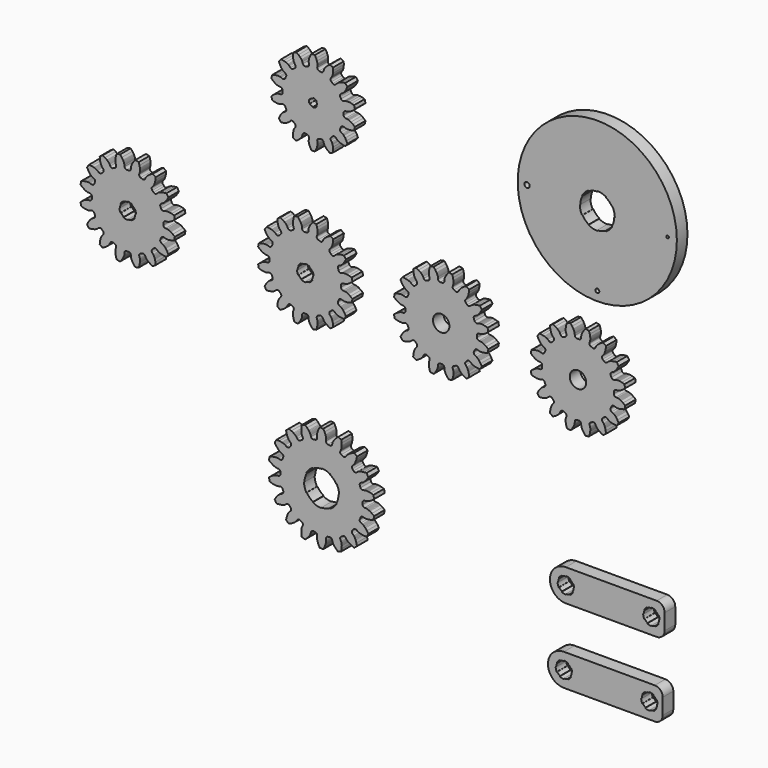
from build123d import *

# Parameters (mm, degrees)
F1_DEPTH = 5
F0_R     = 3.1
F0_R_2   = 30
F0_R_3   = 0.75
F0_R_4   = 1
F0_R_5   = 0.5


# Not quite as in the source:
# - ends of sketch curves that miss each other by under 0.0002 mm in the source are joined


with BuildPart() as f1:
    # F0 (on Front) → F1 (new body)
    with BuildSketch(Plane.XZ):
        with BuildLine():
            ThreePointArc((-63.9951395741, 71.3684795882), (-64.546172127, 71.1185368), (-65.1191699867, 71.3129120157))
            ThreePointArc((-65.1191699867, 71.3129120157), (-65.3881380938, 71.534151901), (-65.6636821129, 71.7471458493))
            ThreePointArc((-65.6636821129, 71.7471458493), (-65.9806878227, 72.2625256994), (-65.8596280407, 72.8553600266))
            Line((-65.8596280407, 72.8553600266), (-65.538945, 73.348971))
            Line((-65.538945, 73.348971), (-65.378251, 73.602757))
            Line((-65.378251, 73.602757), (-65.330022, 73.699631))
            Line((-65.330022, 73.699631), (-65.272467, 73.836879))
            Line((-65.272467, 73.836879), (-65.215385, 73.998994))
            Line((-65.215385, 73.998994), (-65.039238, 74.804267))
            Line((-65.039238, 74.804267), (-64.981947, 75.684169))
            Line((-64.981947, 75.684169), (-65.04075, 76.667073))
            ThreePointArc((-65.04075, 76.667073), (-65.616130958, 76.9585917824), (-66.2027938918, 77.2266832499))
            Line((-66.2027938918, 77.2266832499), (-67.007923, 76.659828))
            Line((-67.007923, 76.659828), (-67.660137, 76.066426))
            Line((-67.660137, 76.066426), (-68.179899, 75.426629))
            Line((-68.179899, 75.426629), (-68.271056, 75.280923))
            Line((-68.271056, 75.280923), (-68.342475, 75.150352))
            Line((-68.342475, 75.150352), (-68.388144, 75.052245))
            Line((-68.388144, 75.052245), (-68.486371, 74.768377))
            Line((-68.486371, 74.768377), (-68.672349, 74.209894))
            ThreePointArc((-68.672349, 74.209894), (-69.0603667079, 73.7456198609), (-69.6609560474, 73.6721318179))
            ThreePointArc((-69.6609560474, 73.6721318179), (-69.999280113, 73.7547609566), (-70.339951049, 73.8271077506))
            ThreePointArc((-70.339951049, 73.8271077506), (-70.8491783878, 74.1539045989), (-70.9973289409, 74.7405559923))
            Line((-70.9973289409, 74.7405559923), (-70.922573, 75.324424))
            Line((-70.922573, 75.324424), (-70.887906, 75.622799))
            Line((-70.887906, 75.622799), (-70.886486, 75.731006))
            Line((-70.886486, 75.731006), (-70.89418, 75.879634))
            Line((-70.89418, 75.879634), (-70.91309, 76.050462))
            Line((-70.91309, 76.050462), (-71.103781, 76.852415))
            Line((-71.103781, 76.852415), (-71.433939, 77.670037))
            Line((-71.433939, 77.670037), (-71.913385, 78.530089))
            ThreePointArc((-71.913385, 78.530089), (-72.558271, 78.54309), (-73.2031569811, 78.5300885323))
            Line((-73.2031569811, 78.5300885323), (-73.682603, 77.670037))
            Line((-73.682603, 77.670037), (-74.012761, 76.852415))
            Line((-74.012761, 76.852415), (-74.203452, 76.050462))
            Line((-74.203452, 76.050462), (-74.222362, 75.879634))
            Line((-74.222362, 75.879634), (-74.230056, 75.731006))
            Line((-74.230056, 75.731006), (-74.228636, 75.622799))
            Line((-74.228636, 75.622799), (-74.193969, 75.324424))
            Line((-74.193969, 75.324424), (-74.119213, 74.740556))
            ThreePointArc((-74.119213, 74.740556), (-74.2673636122, 74.1539045989), (-74.7765910459, 73.8271082334))
            ThreePointArc((-74.7765910459, 73.8271082334), (-75.117261887, 73.7547609566), (-75.4555858899, 73.6721315773))
            ThreePointArc((-75.4555858899, 73.6721315773), (-76.0561752921, 73.7456198609), (-76.4441926358, 74.2098941206))
            Line((-76.4441926358, 74.2098941206), (-76.630171, 74.768377))
            Line((-76.630171, 74.768377), (-76.728398, 75.052245))
            Line((-76.728398, 75.052245), (-76.774067, 75.150352))
            Line((-76.774067, 75.150352), (-76.845486, 75.280923))
            Line((-76.845486, 75.280923), (-76.936643, 75.426629))
            Line((-76.936643, 75.426629), (-77.456405, 76.066426))
            Line((-77.456405, 76.066426), (-78.108619, 76.659828))
            Line((-78.108619, 76.659828), (-78.913748, 77.226683))
            ThreePointArc((-78.913748, 77.226683), (-79.500411042, 76.9585917824), (-80.0757917391, 76.6670725098))
            Line((-80.0757917391, 76.6670725098), (-80.134595, 75.684169))
            Line((-80.134595, 75.684169), (-80.077304, 74.804267))
            Line((-80.077304, 74.804267), (-79.901157, 73.998994))
            Line((-79.901157, 73.998994), (-79.844075, 73.836879))
            Line((-79.844075, 73.836879), (-79.78652, 73.699631))
            Line((-79.78652, 73.699631), (-79.738291, 73.602757))
            Line((-79.738291, 73.602757), (-79.577597, 73.348971))
            Line((-79.577597, 73.348971), (-79.256913, 72.85536))
            ThreePointArc((-79.256913, 72.85536), (-79.1358541773, 72.2625256994), (-79.4528598452, 71.7471467934))
            ThreePointArc((-79.4528598452, 71.7471467934), (-79.7284039062, 71.534151901), (-79.997371955, 71.312911947))
            ThreePointArc((-79.997371955, 71.312911947), (-80.570369873, 71.1185368), (-81.1214024259, 71.3684795882))
            Line((-81.1214024259, 71.3684795882), (-81.531279, 71.790962))
            Line((-81.531279, 71.790962), (-81.742944, 72.004099))
            Line((-81.742944, 72.004099), (-81.826658, 72.072675))
            Line((-81.826658, 72.072675), (-81.947657, 72.159328))
            Line((-81.947657, 72.159328), (-82.093006, 72.251053))
            Line((-82.093006, 72.251053), (-82.838892, 72.601974))
            Line((-82.838892, 72.601974), (-83.683985, 72.853625))
            Line((-83.683985, 72.853625), (-84.65533, 73.015013))
            ThreePointArc((-84.65533, 73.015013), (-85.0675744009, 72.5189272292), (-85.4594890935, 72.0066290686))
            Line((-85.4594890935, 72.0066290686), (-85.086004, 71.095549))
            Line((-85.086004, 71.095549), (-84.652611, 70.327642))
            Line((-84.652611, 70.327642), (-84.144513, 69.678544))
            Line((-84.144513, 69.678544), (-84.022745, 69.55725))
            Line((-84.022745, 69.55725), (-83.91134, 69.458567))
            Line((-83.91134, 69.458567), (-83.825855, 69.392212))
            Line((-83.825855, 69.392212), (-83.570962, 69.233281))
            Line((-83.570962, 69.233281), (-83.067865, 68.927692))
            ThreePointArc((-83.067865, 68.927692), (-82.7015732777, 68.4460920126), (-82.7635712642, 67.8442081373))
            ThreePointArc((-82.7635712642, 67.8442081373), (-82.9194129075, 67.5327531522), (-83.0657522766, 67.216722123))
            ThreePointArc((-83.0657522766, 67.216722123), (-83.497669733, 66.7929815097), (-84.1025789525, 66.7790881289))
            Line((-84.1025789525, 66.7790881289), (-84.655173, 66.981892))
            Line((-84.655173, 66.981892), (-84.938354, 67.082084))
            Line((-84.938354, 67.082084), (-85.043531, 67.107547))
            Line((-85.043531, 67.107547), (-85.190145, 67.133119))
            Line((-85.190145, 67.133119), (-85.360897, 67.152696))
            Line((-85.360897, 67.152696), (-86.185177, 67.145237))
            Line((-86.185177, 67.145237), (-87.055767, 67.005295))
            Line((-87.055767, 67.005295), (-88.000942, 66.729249))
            ThreePointArc((-88.000942, 66.729249), (-88.1571175814, 66.1034250025), (-88.2879426512, 65.4718149351))
            Line((-88.2879426512, 65.4718149351), (-87.556141, 64.81301))
            Line((-87.556141, 64.81301), (-86.832486, 64.309192))
            Line((-86.832486, 64.309192), (-86.093072, 63.94483))
            Line((-86.093072, 63.94483), (-85.930735, 63.888381))
            Line((-85.930735, 63.888381), (-85.787546, 63.847807))
            Line((-85.787546, 63.847807), (-85.681736, 63.825114))
            Line((-85.681736, 63.825114), (-85.383128, 63.792517))
            Line((-85.383128, 63.792517), (-84.797263, 63.735476))
            ThreePointArc((-84.797263, 63.735476), (-84.2582864927, 63.4604974264), (-84.052997411, 62.8913180125))
            ThreePointArc((-84.052997411, 62.8913180125), (-84.058271, 62.54309), (-84.0529974983, 62.1948620152))
            ThreePointArc((-84.0529974983, 62.1948620152), (-84.2582864927, 61.6256825736), (-84.7972630169, 61.3507041768))
            Line((-84.7972630169, 61.3507041768), (-85.383128, 61.293663))
            Line((-85.383128, 61.293663), (-85.681736, 61.261066))
            Line((-85.681736, 61.261066), (-85.787546, 61.238373))
            Line((-85.787546, 61.238373), (-85.930735, 61.197799))
            Line((-85.930735, 61.197799), (-86.093072, 61.14135))
            Line((-86.093072, 61.14135), (-86.832486, 60.776988))
            Line((-86.832486, 60.776988), (-87.556141, 60.27317))
            Line((-87.556141, 60.27317), (-88.287943, 59.614365))
            ThreePointArc((-88.287943, 59.614365), (-88.1571175814, 58.9827549975), (-88.000941554, 58.3569311209))
            Line((-88.000941554, 58.3569311209), (-87.055767, 58.080885))
            Line((-87.055767, 58.080885), (-86.185177, 57.940943))
            Line((-86.185177, 57.940943), (-85.360897, 57.933484))
            Line((-85.360897, 57.933484), (-85.190145, 57.953061))
            Line((-85.190145, 57.953061), (-85.043531, 57.978633))
            Line((-85.043531, 57.978633), (-84.938354, 58.004096))
            Line((-84.938354, 58.004096), (-84.655173, 58.104288))
            Line((-84.655173, 58.104288), (-84.102579, 58.307093))
            ThreePointArc((-84.102579, 58.307093), (-83.497669733, 58.2931984903), (-83.0657527485, 57.8694581119))
            ThreePointArc((-83.0657527485, 57.8694581119), (-82.9194129075, 57.5534268478), (-82.7635709946, 57.2419720028))
            ThreePointArc((-82.7635709946, 57.2419720028), (-82.7015732077, 56.6400882366), (-83.0678648177, 56.1584886987))
            Line((-83.0678648177, 56.1584886987), (-83.570962, 55.852899))
            Line((-83.570962, 55.852899), (-83.825855, 55.693968))
            Line((-83.825855, 55.693968), (-83.91134, 55.627613))
            Line((-83.91134, 55.627613), (-84.022745, 55.52893))
            Line((-84.022745, 55.52893), (-84.144513, 55.407636))
            Line((-84.144513, 55.407636), (-84.652611, 54.758538))
            Line((-84.652611, 54.758538), (-85.086004, 53.990631))
            Line((-85.086004, 53.990631), (-85.459489, 53.079551))
            ThreePointArc((-85.459489, 53.079551), (-85.0675744009, 52.5672527708), (-84.6553298165, 52.0711671589))
            Line((-84.6553298165, 52.0711671589), (-83.683985, 52.232555))
            Line((-83.683985, 52.232555), (-82.838892, 52.484206))
            Line((-82.838892, 52.484206), (-82.093006, 52.835127))
            Line((-82.093006, 52.835127), (-81.947657, 52.926852))
            Line((-81.947657, 52.926852), (-81.826658, 53.013505))
            Line((-81.826658, 53.013505), (-81.742944, 53.082081))
            Line((-81.742944, 53.082081), (-81.531279, 53.295218))
            Line((-81.531279, 53.295218), (-81.121403, 53.717701))
            ThreePointArc((-81.121403, 53.717701), (-80.570369514, 53.9676432178), (-79.9973720133, 53.7732679843))
            ThreePointArc((-79.9973720133, 53.7732679843), (-79.7284039062, 53.552028099), (-79.4528598871, 53.3390341507))
            ThreePointArc((-79.4528598871, 53.3390341507), (-79.1358543024, 52.8236550082), (-79.2569135017, 52.230820675))
            Line((-79.2569135017, 52.230820675), (-79.577597, 51.737209))
            Line((-79.577597, 51.737209), (-79.738291, 51.483423))
            Line((-79.738291, 51.483423), (-79.78652, 51.386549))
            Line((-79.78652, 51.386549), (-79.844075, 51.249301))
            Line((-79.844075, 51.249301), (-79.901157, 51.087186))
            Line((-79.901157, 51.087186), (-80.077304, 50.281913))
            Line((-80.077304, 50.281913), (-80.134595, 49.402011))
            Line((-80.134595, 49.402011), (-80.075792, 48.419107))
            ThreePointArc((-80.075792, 48.419107), (-79.5004112536, 48.1275883196), (-78.9137481082, 47.8594967501))
            Line((-78.9137481082, 47.8594967501), (-78.108619, 48.426352))
            Line((-78.108619, 48.426352), (-77.456405, 49.019754))
            Line((-77.456405, 49.019754), (-76.936643, 49.659551))
            Line((-76.936643, 49.659551), (-76.845486, 49.805257))
            Line((-76.845486, 49.805257), (-76.774067, 49.935828))
            Line((-76.774067, 49.935828), (-76.728398, 50.033935))
            Line((-76.728398, 50.033935), (-76.630171, 50.317803))
            Line((-76.630171, 50.317803), (-76.444193, 50.876286))
            ThreePointArc((-76.444193, 50.876286), (-76.0561752921, 51.3405601391), (-75.4555859526, 51.4140481821))
            ThreePointArc((-75.4555859526, 51.4140481821), (-75.1172620099, 51.3314190714), (-74.776590951, 51.2590722494))
            ThreePointArc((-74.776590951, 51.2590722494), (-74.2673636122, 50.9322754011), (-74.1192130591, 50.3456240077))
            Line((-74.1192130591, 50.3456240077), (-74.193969, 49.761756))
            Line((-74.193969, 49.761756), (-74.228636, 49.463381))
            Line((-74.228636, 49.463381), (-74.230056, 49.355174))
            Line((-74.230056, 49.355174), (-74.222362, 49.206546))
            Line((-74.222362, 49.206546), (-74.203452, 49.035718))
            Line((-74.203452, 49.035718), (-74.012761, 48.233765))
            Line((-74.012761, 48.233765), (-73.682603, 47.416143))
            Line((-73.682603, 47.416143), (-73.203157, 46.556091))
            ThreePointArc((-73.203157, 46.556091), (-72.558271, 46.54309), (-71.9133849786, 46.5560914693))
            Line((-71.9133849786, 46.5560914693), (-71.433939, 47.416143))
            Line((-71.433939, 47.416143), (-71.103781, 48.233765))
            Line((-71.103781, 48.233765), (-70.91309, 49.035718))
            Line((-70.91309, 49.035718), (-70.89418, 49.206546))
            Line((-70.89418, 49.206546), (-70.886486, 49.355174))
            Line((-70.886486, 49.355174), (-70.887906, 49.463381))
            Line((-70.887906, 49.463381), (-70.922573, 49.761756))
            Line((-70.922573, 49.761756), (-70.997329, 50.345624))
            ThreePointArc((-70.997329, 50.345624), (-70.8491783878, 50.9322754011), (-70.3399509541, 51.2590717666))
            ThreePointArc((-70.3399509541, 51.2590717666), (-69.9992799901, 51.3314190714), (-69.6609558662, 51.4140484862))
            ThreePointArc((-69.6609558662, 51.4140484862), (-69.0603667079, 51.3405601391), (-68.6723493642, 50.8762858794))
            Line((-68.6723493642, 50.8762858794), (-68.486371, 50.317803))
            Line((-68.486371, 50.317803), (-68.388144, 50.033935))
            Line((-68.388144, 50.033935), (-68.342475, 49.935828))
            Line((-68.342475, 49.935828), (-68.271056, 49.805257))
            Line((-68.271056, 49.805257), (-68.179899, 49.659551))
            Line((-68.179899, 49.659551), (-67.660137, 49.019754))
            Line((-67.660137, 49.019754), (-67.007923, 48.426352))
            Line((-67.007923, 48.426352), (-66.202794, 47.859497))
            ThreePointArc((-66.202794, 47.859497), (-65.6161307464, 48.1275883196), (-65.0407498462, 48.4191077109))
            Line((-65.0407498462, 48.4191077109), (-64.981947, 49.402011))
            Line((-64.981947, 49.402011), (-65.039238, 50.281913))
            Line((-65.039238, 50.281913), (-65.215385, 51.087186))
            Line((-65.215385, 51.087186), (-65.272467, 51.249301))
            Line((-65.272467, 51.249301), (-65.330022, 51.386549))
            Line((-65.330022, 51.386549), (-65.378251, 51.483423))
            Line((-65.378251, 51.483423), (-65.538945, 51.737209))
            Line((-65.538945, 51.737209), (-65.859629, 52.23082))
            ThreePointArc((-65.859629, 52.23082), (-65.9806876976, 52.8236550082), (-65.6636816749, 53.339033566))
            ThreePointArc((-65.6636816749, 53.339033566), (-65.3881380938, 53.552028099), (-65.119170045, 53.773268053))
            ThreePointArc((-65.119170045, 53.773268053), (-64.546172486, 53.9676432178), (-63.9951400738, 53.7177009287))
            Line((-63.9951400738, 53.7177009287), (-63.585263, 53.295218))
            Line((-63.585263, 53.295218), (-63.373598, 53.082081))
            Line((-63.373598, 53.082081), (-63.289884, 53.013505))
            Line((-63.289884, 53.013505), (-63.168885, 52.926852))
            Line((-63.168885, 52.926852), (-63.023536, 52.835127))
            Line((-63.023536, 52.835127), (-62.27765, 52.484206))
            Line((-62.27765, 52.484206), (-61.432557, 52.232555))
            Line((-61.432557, 52.232555), (-60.461212, 52.071167))
            ThreePointArc((-60.461212, 52.071167), (-60.0489675991, 52.5672527708), (-59.6570529065, 53.0795509314))
            Line((-59.6570529065, 53.0795509314), (-60.030538, 53.990631))
            Line((-60.030538, 53.990631), (-60.463931, 54.758538))
            Line((-60.463931, 54.758538), (-60.972029, 55.407636))
            Line((-60.972029, 55.407636), (-61.093797, 55.52893))
            Line((-61.093797, 55.52893), (-61.205202, 55.627613))
            Line((-61.205202, 55.627613), (-61.290687, 55.693968))
            Line((-61.290687, 55.693968), (-61.54558, 55.852899))
            Line((-61.54558, 55.852899), (-62.048677, 56.158488))
            ThreePointArc((-62.048677, 56.158488), (-62.4149687923, 56.6400882366), (-62.3529707358, 57.2419718627))
            ThreePointArc((-62.3529707358, 57.2419718627), (-62.1971290925, 57.5534268478), (-62.0507897234, 57.869457877))
            ThreePointArc((-62.0507897234, 57.869457877), (-61.618872267, 58.2931984903), (-61.0139630475, 58.3070918711))
            Line((-61.0139630475, 58.3070918711), (-60.461369, 58.104288))
            Line((-60.461369, 58.104288), (-60.178188, 58.004096))
            Line((-60.178188, 58.004096), (-60.073011, 57.978633))
            Line((-60.073011, 57.978633), (-59.926397, 57.953061))
            Line((-59.926397, 57.953061), (-59.755645, 57.933484))
            Line((-59.755645, 57.933484), (-58.931365, 57.940943))
            Line((-58.931365, 57.940943), (-58.060775, 58.080885))
            Line((-58.060775, 58.080885), (-57.1156, 58.356931))
            ThreePointArc((-57.1156, 58.356931), (-56.9594244186, 58.9827549975), (-56.8285993488, 59.6143650649))
            Line((-56.8285993488, 59.6143650649), (-57.560401, 60.27317))
            Line((-57.560401, 60.27317), (-58.284056, 60.776988))
            Line((-58.284056, 60.776988), (-59.02347, 61.14135))
            Line((-59.02347, 61.14135), (-59.185807, 61.197799))
            Line((-59.185807, 61.197799), (-59.328996, 61.238373))
            Line((-59.328996, 61.238373), (-59.434806, 61.261066))
            Line((-59.434806, 61.261066), (-59.733414, 61.293663))
            Line((-59.733414, 61.293663), (-60.319279, 61.350704))
            ThreePointArc((-60.319279, 61.350704), (-60.8582555073, 61.6256825736), (-61.063544589, 62.1948619875))
            ThreePointArc((-61.063544589, 62.1948619875), (-61.058271, 62.54309), (-61.0635445026, 62.8913180151))
            ThreePointArc((-61.0635445026, 62.8913180151), (-60.8582555073, 63.4604974264), (-60.3192789831, 63.7354758232))
            Line((-60.3192789831, 63.7354758232), (-59.733414, 63.792517))
            Line((-59.733414, 63.792517), (-59.434806, 63.825114))
            Line((-59.434806, 63.825114), (-59.328996, 63.847807))
            Line((-59.328996, 63.847807), (-59.185807, 63.888381))
            Line((-59.185807, 63.888381), (-59.02347, 63.94483))
            Line((-59.02347, 63.94483), (-58.284056, 64.309192))
            Line((-58.284056, 64.309192), (-57.560401, 64.81301))
            Line((-57.560401, 64.81301), (-56.828599, 65.471815))
            ThreePointArc((-56.828599, 65.471815), (-56.9594244186, 66.1034250025), (-57.115600446, 66.7292488791))
            Line((-57.115600446, 66.7292488791), (-58.060775, 67.005295))
            Line((-58.060775, 67.005295), (-58.931365, 67.145237))
            Line((-58.931365, 67.145237), (-59.755645, 67.152696))
            Line((-59.755645, 67.152696), (-59.926397, 67.133119))
            Line((-59.926397, 67.133119), (-60.073011, 67.107547))
            Line((-60.073011, 67.107547), (-60.178188, 67.082084))
            Line((-60.178188, 67.082084), (-60.461369, 66.981892))
            Line((-60.461369, 66.981892), (-61.013963, 66.779087))
            ThreePointArc((-61.013963, 66.779087), (-61.618872267, 66.7929815097), (-62.0507892515, 67.2167218881))
            ThreePointArc((-62.0507892515, 67.2167218881), (-62.1971290925, 67.5327531522), (-62.3529710054, 67.8442079972))
            ThreePointArc((-62.3529710054, 67.8442079972), (-62.4149687223, 68.4460920126), (-62.0486767394, 68.9276915693))
            Line((-62.0486767394, 68.9276915693), (-61.54558, 69.233281))
            Line((-61.54558, 69.233281), (-61.290687, 69.392212))
            Line((-61.290687, 69.392212), (-61.205202, 69.458567))
            Line((-61.205202, 69.458567), (-61.093797, 69.55725))
            Line((-61.093797, 69.55725), (-60.972029, 69.678544))
            Line((-60.972029, 69.678544), (-60.463931, 70.327642))
            Line((-60.463931, 70.327642), (-60.030538, 71.095549))
            Line((-60.030538, 71.095549), (-59.657053, 72.006629))
            ThreePointArc((-59.657053, 72.006629), (-60.0489675991, 72.5189272292), (-60.4612121835, 73.0150128411))
            Line((-60.4612121835, 73.0150128411), (-61.432557, 72.853625))
            Line((-61.432557, 72.853625), (-62.27765, 72.601974))
            Line((-62.27765, 72.601974), (-63.023536, 72.251053))
            Line((-63.023536, 72.251053), (-63.168885, 72.159328))
            Line((-63.168885, 72.159328), (-63.289884, 72.072675))
            Line((-63.289884, 72.072675), (-63.373598, 72.004099))
            Line((-63.373598, 72.004099), (-63.585263, 71.790962))
            Line((-63.585263, 71.790962), (-63.9951395741, 71.3684795882))
        make_face()
        with BuildLine():
            ThreePointArc((-73.770706674, 63.2430898118), (-73.2582710941, 63.755525511), (-72.558271, 63.94309))
            Line((-72.558271, 63.94309), (-72.558271, 64.14309))
            ThreePointArc((-72.558271, 64.14309), (-71.7582709234, 63.9287306018), (-71.1726302655, 63.3430898467))
            Line((-71.1726302655, 63.3430898467), (-71.345835, 63.24309))
            ThreePointArc((-71.345835, 63.24309), (-71.158271, 62.54309), (-71.345835326, 61.8430901882))
            Line((-71.345835326, 61.8430901882), (-71.17263, 61.74309))
            ThreePointArc((-71.17263, 61.74309), (-71.7582709234, 61.1574493982), (-72.558271, 60.94309))
            Line((-72.558271, 60.94309), (-72.558271, 61.14309))
            ThreePointArc((-72.558271, 61.14309), (-73.2582710941, 61.330654489), (-73.770706674, 61.8430901882))
            Line((-73.770706674, 61.8430901882), (-73.943912, 61.74309))
            ThreePointArc((-73.943912, 61.74309), (-74.158271, 62.54309), (-73.9439117345, 63.3430898467))
            Line((-73.9439117345, 63.3430898467), (-73.770706674, 63.2430898118))
        make_face(mode=Mode.SUBTRACT)
    extrude(amount=F1_DEPTH)


with BuildPart() as f1b:
    # F0 (on Front) → F1, piece 2 (new body)
    with BuildSketch(Plane.XZ):
        with BuildLine():
            Line((-70.960719, -82.299435), (-70.87534, -82.592835))
            Line((-70.87534, -82.592835), (-70.542866, -83.456846))
            Line((-70.542866, -83.456846), (-70.067808, -84.371709))
            ThreePointArc((-70.067808, -84.371709), (-69.387823, -84.383272), (-68.7078379943, -84.3717091673))
            Line((-68.7078379943, -84.3717091673), (-68.23278, -83.456846))
            Line((-68.23278, -83.456846), (-67.900306, -82.592835))
            Line((-67.900306, -82.592835), (-67.814927, -82.299435))
            Line((-67.814927, -82.299435), (-67.748498, -82.021591))
            Line((-67.748498, -82.021591), (-67.700855, -81.763606))
            Line((-67.700855, -81.763606), (-67.671642, -81.531442))
            Line((-67.671642, -81.531442), (-67.6603, -81.332169))
            Line((-67.6603, -81.332169), (-67.667666, -81.151475))
            Line((-67.667666, -81.151475), (-67.724501, -80.583157))
            ThreePointArc((-67.724501, -80.583157), (-67.5611978841, -80.0086093638), (-67.0465579891, -79.7054280712))
            ThreePointArc((-67.0465579891, -79.7054280712), (-66.6962760548, -79.6477921379), (-66.3474059848, -79.5821490761))
            ThreePointArc((-66.3474059848, -79.5821490761), (-65.7601091451, -79.691028895), (-65.4101468966, -80.1750729741))
            Line((-65.4101468966, -80.1750729741), (-65.269178, -80.728557))
            Line((-65.269178, -80.728557), (-65.214299, -80.900873))
            Line((-65.214299, -80.900873), (-65.135486, -81.084249))
            Line((-65.135486, -81.084249), (-65.02863, -81.292421))
            Line((-65.02863, -81.292421), (-64.895624, -81.518552))
            Line((-64.895624, -81.518552), (-64.738173, -81.75692))
            Line((-64.738173, -81.75692), (-64.557594, -82.003425))
            Line((-64.557594, -82.003425), (-63.949661, -82.701617))
            Line((-63.949661, -82.701617), (-63.190351, -83.398827))
            ThreePointArc((-63.190351, -83.398827), (-62.5474201228, -83.1771244118), (-61.9123987379, -82.9336906503))
            Line((-61.9123987379, -82.9336906503), (-61.778892, -81.911521))
            Line((-61.778892, -81.911521), (-61.761977, -80.985903))
            Line((-61.761977, -80.985903), (-61.782096, -80.680996))
            Line((-61.782096, -80.680996), (-61.814701, -80.397188))
            Line((-61.814701, -80.397188), (-61.858168, -80.138467))
            Line((-61.858168, -80.138467), (-61.910121, -79.910312))
            Line((-61.910121, -79.910312), (-61.967618, -79.719178))
            Line((-61.967618, -79.719178), (-62.036341, -79.551901))
            Line((-62.036341, -79.551901), (-62.284125, -79.037295))
            ThreePointArc((-62.284125, -79.037295), (-62.3271768832, -78.441543438), (-61.9472676129, -77.9806287075))
            ThreePointArc((-61.9472676129, -77.9806287075), (-61.6378228438, -77.8066656684), (-61.3324439541, -77.6256610755))
            ThreePointArc((-61.3324439541, -77.6256610755), (-60.7433260438, -77.5271065635), (-60.2489159887, -77.8622649924))
            Line((-60.2489159887, -77.8622649924), (-59.927146, -78.334156))
            Line((-59.927146, -78.334156), (-59.816641, -78.477311))
            Line((-59.816641, -78.477311), (-59.679862, -78.622672))
            Line((-59.679862, -78.622672), (-59.508252, -78.781742))
            Line((-59.508252, -78.781742), (-59.305926, -78.948746))
            Line((-59.305926, -78.948746), (-59.076444, -79.118887))
            Line((-59.076444, -79.118887), (-58.822445, -79.288764))
            Line((-58.822445, -79.288764), (-58.01238, -79.736924))
            Line((-58.01238, -79.736924), (-57.060402, -80.132389))
            ThreePointArc((-57.060402, -80.132389), (-56.532070839, -79.7041608898), (-56.0186046438, -79.2582173963))
            Line((-56.0186046438, -79.2582173963), (-56.242752, -78.25203))
            Line((-56.242752, -78.25203), (-56.543438, -77.376449))
            Line((-56.543438, -77.376449), (-56.666627, -77.096811))
            Line((-56.666627, -77.096811), (-56.794334, -76.841271))
            Line((-56.794334, -76.841271), (-56.923667, -76.613018))
            Line((-56.923667, -76.613018), (-57.050521, -76.416393))
            Line((-57.050521, -76.416393), (-57.169922, -76.25645))
            Line((-57.169922, -76.25645), (-57.291713, -76.122766))
            Line((-57.291713, -76.122766), (-57.700559, -75.723941))
            ThreePointArc((-57.700559, -75.723941), (-57.9447733652, -75.1788424208), (-57.7454175578, -74.6157883887))
            ThreePointArc((-57.7454175578, -74.6157883887), (-57.5141342851, -74.346480133), (-57.2890787703, -74.0719451839))
            ThreePointArc((-57.2890787703, -74.0719451839), (-56.7691964636, -73.7778445262), (-56.1899724403, -73.9236926072))
            Line((-56.1899724403, -73.9236926072), (-55.726211, -74.257073))
            Line((-55.726211, -74.257073), (-55.573409, -74.3538))
            Line((-55.573409, -74.3538), (-55.395163, -74.443613))
            Line((-55.395163, -74.443613), (-55.179496, -74.534396))
            Line((-55.179496, -74.534396), (-54.932253, -74.622128))
            Line((-54.932253, -74.622128), (-54.658419, -74.703521))
            Line((-54.658419, -74.703521), (-54.361637, -74.776281))
            Line((-54.361637, -74.776281), (-53.447145, -74.920355))
            Line((-53.447145, -74.920355), (-52.417321, -74.966374))
            ThreePointArc((-52.417321, -74.966374), (-52.0673147589, -74.3832717136), (-51.7373361988, -73.7886064269))
            Line((-51.7373361988, -73.7886064269), (-52.292102, -72.919763))
            Line((-52.292102, -72.919763), (-52.874121, -72.199826))
            Line((-52.874121, -72.199826), (-53.085523, -71.979185))
            Line((-53.085523, -71.979185), (-53.292928, -71.782735))
            Line((-53.292928, -71.782735), (-53.492528, -71.612482))
            Line((-53.492528, -71.612482), (-53.678982, -71.471101))
            Line((-53.678982, -71.471101), (-53.845886, -71.361642))
            Line((-53.845886, -71.361642), (-54.006055, -71.277674))
            Line((-54.006055, -71.277674), (-54.52665, -71.042736))
            ThreePointArc((-54.52665, -71.042736), (-54.9425715037, -70.6140368055), (-54.9478140305, -70.0167543783))
            ThreePointArc((-54.9478140305, -70.0167543783), (-54.8225872783, -69.6845839481), (-54.7050008024, -69.3496320668))
            ThreePointArc((-54.7050008024, -69.3496320668), (-54.31706012, -68.8954580934), (-53.7228841047, -68.8344043664))
            Line((-53.7228841047, -68.8344043664), (-53.173069, -68.989064))
            Line((-53.173069, -68.989064), (-52.996399, -69.027695))
            Line((-52.996399, -69.027695), (-52.798184, -69.051128))
            Line((-52.798184, -69.051128), (-52.564474, -69.062674))
            Line((-52.564474, -69.062674), (-52.302135, -69.060554))
            Line((-52.302135, -69.060554), (-52.016978, -69.043381))
            Line((-52.016978, -69.043381), (-51.713209, -69.010247))
            Line((-51.713209, -69.010247), (-50.80459, -68.832858))
            Line((-50.80459, -68.832858), (-49.821133, -68.523882))
            ThreePointArc((-49.821133, -68.523882), (-49.6916679224, -67.8562354549), (-49.5849770642, -67.1845739909))
            Line((-49.5849770642, -67.1845739909), (-50.403448, -66.557869))
            Line((-50.403448, -66.557869), (-51.1966, -66.080412))
            Line((-51.1966, -66.080412), (-51.470717, -65.945381))
            Line((-51.470717, -65.945381), (-51.732804, -65.831714))
            Line((-51.732804, -65.831714), (-51.978596, -65.739997))
            Line((-51.978596, -65.739997), (-52.202161, -65.670913))
            Line((-52.202161, -65.670913), (-52.396436, -65.625139))
            Line((-52.396436, -65.625139), (-52.575664, -65.601016))
            Line((-52.575664, -65.601016), (-53.145218, -65.5583))
            ThreePointArc((-53.145218, -65.5583), (-53.6826793906, -65.2977082395), (-53.891888223, -64.7382400178))
            ThreePointArc((-53.891888223, -64.7382400178), (-53.887823, -64.383272), (-53.8918881227, -64.0283040028))
            ThreePointArc((-53.8918881227, -64.0283040028), (-53.6826793668, -63.4688357344), (-53.1452179637, -63.2082435129))
            Line((-53.1452179637, -63.2082435129), (-52.575664, -63.165528))
            Line((-52.575664, -63.165528), (-52.396436, -63.141405))
            Line((-52.396436, -63.141405), (-52.202161, -63.095631))
            Line((-52.202161, -63.095631), (-51.978596, -63.026547))
            Line((-51.978596, -63.026547), (-51.732804, -62.93483))
            Line((-51.732804, -62.93483), (-51.470717, -62.821163))
            Line((-51.470717, -62.821163), (-51.1966, -62.686132))
            Line((-51.1966, -62.686132), (-50.403448, -62.208675))
            Line((-50.403448, -62.208675), (-49.584977, -61.58197))
            ThreePointArc((-49.584977, -61.58197), (-49.6916680073, -60.9103080633), (-49.8211332563, -60.2426618426))
            Line((-49.8211332563, -60.2426618426), (-50.80459, -59.933686))
            Line((-50.80459, -59.933686), (-51.713209, -59.756297))
            Line((-51.713209, -59.756297), (-52.016978, -59.723163))
            Line((-52.016978, -59.723163), (-52.302135, -59.70599))
            Line((-52.302135, -59.70599), (-52.564474, -59.70387))
            Line((-52.564474, -59.70387), (-52.798184, -59.715416))
            Line((-52.798184, -59.715416), (-52.996399, -59.738849))
            Line((-52.996399, -59.738849), (-53.173069, -59.77748))
            Line((-53.173069, -59.77748), (-53.722884, -59.932139))
            ThreePointArc((-53.722884, -59.932139), (-54.3170604178, -59.8710857504), (-54.7050019944, -59.4169109981))
            ThreePointArc((-54.7050019944, -59.4169109981), (-54.8225875996, -59.0819591692), (-54.947814057, -58.7497880223))
            ThreePointArc((-54.947814057, -58.7497880223), (-54.9425712495, -58.1525065751), (-54.5266497062, -57.7238076584))
            Line((-54.5266497062, -57.7238076584), (-54.006055, -57.48887))
            Line((-54.006055, -57.48887), (-53.845886, -57.404902))
            Line((-53.845886, -57.404902), (-53.678982, -57.295443))
            Line((-53.678982, -57.295443), (-53.492528, -57.154062))
            Line((-53.492528, -57.154062), (-53.292928, -56.983809))
            Line((-53.292928, -56.983809), (-53.085523, -56.787359))
            Line((-53.085523, -56.787359), (-52.874121, -56.566718))
            Line((-52.874121, -56.566718), (-52.292102, -55.846781))
            Line((-52.292102, -55.846781), (-51.7373366139, -54.9779367942))
            ThreePointArc((-51.7373366139, -54.9779367942), (-52.0673151917, -54.3832715369), (-52.4173211536, -53.8001690958))
            Line((-52.4173211536, -53.8001690958), (-53.447145, -53.846189))
            Line((-53.447145, -53.846189), (-54.361637, -53.990263))
            Line((-54.361637, -53.990263), (-54.658419, -54.063023))
            Line((-54.658419, -54.063023), (-54.932253, -54.144416))
            Line((-54.932253, -54.144416), (-55.179496, -54.232148))
            Line((-55.179496, -54.232148), (-55.395163, -54.322931))
            Line((-55.395163, -54.322931), (-55.573409, -54.412744))
            Line((-55.573409, -54.412744), (-55.726211, -54.509471))
            Line((-55.726211, -54.509471), (-56.189972, -54.842851))
            ThreePointArc((-56.189972, -54.842851), (-56.7691965595, -54.9886994609), (-57.2890791005, -54.6945990805))
            ThreePointArc((-57.2890791005, -54.6945990805), (-57.5141347774, -54.4200632803), (-57.7454184556, -54.1507544004))
            ThreePointArc((-57.7454184556, -54.1507544004), (-57.9447733359, -53.5877008566), (-57.7005594255, -53.0426025938))
            Line((-57.7005594255, -53.0426025938), (-57.291713, -52.643778))
            Line((-57.291713, -52.643778), (-57.169922, -52.510094))
            Line((-57.169922, -52.510094), (-57.050521, -52.350151))
            Line((-57.050521, -52.350151), (-56.923667, -52.153526))
            Line((-56.923667, -52.153526), (-56.794334, -51.925273))
            Line((-56.794334, -51.925273), (-56.666627, -51.669733))
            Line((-56.666627, -51.669733), (-56.543438, -51.390095))
            Line((-56.543438, -51.390095), (-56.242752, -50.514514))
            Line((-56.242752, -50.514514), (-56.018605, -49.508326))
            ThreePointArc((-56.018605, -49.508326), (-56.5320713311, -49.0623826972), (-57.0604024051, -48.6341545175))
            Line((-57.0604024051, -48.6341545175), (-58.01238, -49.02962))
            Line((-58.01238, -49.02962), (-58.822445, -49.47778))
            Line((-58.822445, -49.47778), (-59.076444, -49.647657))
            Line((-59.076444, -49.647657), (-59.305926, -49.817798))
            Line((-59.305926, -49.817798), (-59.508252, -49.984802))
            Line((-59.508252, -49.984802), (-59.679862, -50.143872))
            Line((-59.679862, -50.143872), (-59.816641, -50.289233))
            Line((-59.816641, -50.289233), (-59.927146, -50.432388))
            Line((-59.927146, -50.432388), (-60.248916, -50.904278))
            ThreePointArc((-60.248916, -50.904278), (-60.743325893, -51.2394374035), (-61.3324441266, -51.1408832082))
            ThreePointArc((-61.3324441266, -51.1408832082), (-61.6378232766, -50.9598780816), (-61.9472672814, -50.7859145142))
            ThreePointArc((-61.9472672814, -50.7859145142), (-62.3271770927, -50.324999905), (-62.2841247165, -49.729248138))
            Line((-62.2841247165, -49.729248138), (-62.036341, -49.214643))
            Line((-62.036341, -49.214643), (-61.967618, -49.047366))
            Line((-61.967618, -49.047366), (-61.910121, -48.856232))
            Line((-61.910121, -48.856232), (-61.858168, -48.628077))
            Line((-61.858168, -48.628077), (-61.814701, -48.369356))
            Line((-61.814701, -48.369356), (-61.782096, -48.085548))
            Line((-61.782096, -48.085548), (-61.761977, -47.780641))
            Line((-61.761977, -47.780641), (-61.778892, -46.855023))
            Line((-61.778892, -46.855023), (-61.912398, -45.832853))
            ThreePointArc((-61.912398, -45.832853), (-62.547420444, -45.5894194712), (-63.1903512261, -45.3677166936))
            Line((-63.1903512261, -45.3677166936), (-63.949661, -46.064927))
            Line((-63.949661, -46.064927), (-64.557594, -46.763119))
            Line((-64.557594, -46.763119), (-64.738173, -47.009624))
            Line((-64.738173, -47.009624), (-64.895624, -47.247992))
            Line((-64.895624, -47.247992), (-65.02863, -47.474123))
            Line((-65.02863, -47.474123), (-65.135486, -47.682295))
            Line((-65.135486, -47.682295), (-65.214299, -47.865671))
            Line((-65.214299, -47.865671), (-65.269178, -48.037987))
            Line((-65.269178, -48.037987), (-65.410147, -48.59147))
            ThreePointArc((-65.410147, -48.59147), (-65.7601088181, -49.0755148981), (-66.347406016, -49.1843950798))
            ThreePointArc((-66.347406016, -49.1843950798), (-66.6962762258, -49.1187518319), (-67.0465580825, -49.06111554))
            ThreePointArc((-67.0465580825, -49.06111554), (-67.5611982343, -48.7579341829), (-67.7245016664, -48.1833860348))
            Line((-67.7245016664, -48.1833860348), (-67.667666, -47.615069))
            Line((-67.667666, -47.615069), (-67.6603, -47.434375))
            Line((-67.6603, -47.434375), (-67.671642, -47.235102))
            Line((-67.671642, -47.235102), (-67.700855, -47.002938))
            Line((-67.700855, -47.002938), (-67.748498, -46.744953))
            Line((-67.748498, -46.744953), (-67.814927, -46.467109))
            Line((-67.814927, -46.467109), (-67.900306, -46.173709))
            Line((-67.900306, -46.173709), (-68.23278, -45.309698))
            Line((-68.23278, -45.309698), (-68.707838, -44.394835))
            ThreePointArc((-68.707838, -44.394835), (-69.387823, -44.383272), (-70.0678079717, -44.3948348315))
            Line((-70.0678079717, -44.3948348315), (-70.542866, -45.309698))
            Line((-70.542866, -45.309698), (-70.87534, -46.173709))
            Line((-70.87534, -46.173709), (-70.960719, -46.467109))
            Line((-70.960719, -46.467109), (-71.027148, -46.744953))
            Line((-71.027148, -46.744953), (-71.074791, -47.002938))
            Line((-71.074791, -47.002938), (-71.104004, -47.235102))
            Line((-71.104004, -47.235102), (-71.115346, -47.434375))
            Line((-71.115346, -47.434375), (-71.10798, -47.615069))
            Line((-71.10798, -47.615069), (-71.051145, -48.183387))
            ThreePointArc((-71.051145, -48.183387), (-71.2144477341, -48.7579341419), (-71.7290878616, -49.061115906))
            ThreePointArc((-71.7290878616, -49.061115906), (-72.0793697742, -49.1187518319), (-72.4282398229, -49.1843948854))
            ThreePointArc((-72.4282398229, -49.1843948854), (-73.0155372845, -49.0755148332), (-73.3654993979, -48.5914698493))
            Line((-73.3654993979, -48.5914698493), (-73.506468, -48.037987))
            Line((-73.506468, -48.037987), (-73.561347, -47.865671))
            Line((-73.561347, -47.865671), (-73.64016, -47.682295))
            Line((-73.64016, -47.682295), (-73.747016, -47.474123))
            Line((-73.747016, -47.474123), (-73.880022, -47.247992))
            Line((-73.880022, -47.247992), (-74.037473, -47.009624))
            Line((-74.037473, -47.009624), (-74.218052, -46.763119))
            Line((-74.218052, -46.763119), (-74.825985, -46.064927))
            Line((-74.825985, -46.064927), (-75.585295, -45.367717))
            ThreePointArc((-75.585295, -45.367717), (-76.2282259918, -45.5894196299), (-76.8632477757, -45.8328535567))
            Line((-76.8632477757, -45.8328535567), (-76.996754, -46.855023))
            Line((-76.996754, -46.855023), (-77.013669, -47.780641))
            Line((-77.013669, -47.780641), (-76.99355, -48.085548))
            Line((-76.99355, -48.085548), (-76.960945, -48.369356))
            Line((-76.960945, -48.369356), (-76.917478, -48.628077))
            Line((-76.917478, -48.628077), (-76.865525, -48.856232))
            Line((-76.865525, -48.856232), (-76.808028, -49.047366))
            Line((-76.808028, -49.047366), (-76.739305, -49.214643))
            Line((-76.739305, -49.214643), (-76.491521, -49.729249))
            ThreePointArc((-76.491521, -49.729249), (-76.4484690406, -50.3250003229), (-76.8283787356, -50.7859154832))
            ThreePointArc((-76.8283787356, -50.7859154832), (-77.1378227234, -50.9598780816), (-77.4432016019, -51.1408826544))
            ThreePointArc((-77.4432016019, -51.1408826544), (-78.0323203805, -51.2394373438), (-78.5267307887, -50.9042778572))
            Line((-78.5267307887, -50.9042778572), (-78.8485, -50.432388))
            Line((-78.8485, -50.432388), (-78.959005, -50.289233))
            Line((-78.959005, -50.289233), (-79.095784, -50.143872))
            Line((-79.095784, -50.143872), (-79.267394, -49.984802))
            Line((-79.267394, -49.984802), (-79.46972, -49.817798))
            Line((-79.46972, -49.817798), (-79.699202, -49.647657))
            Line((-79.699202, -49.647657), (-79.953201, -49.47778))
            Line((-79.953201, -49.47778), (-80.763266, -49.02962))
            Line((-80.763266, -49.02962), (-81.715244, -48.634155))
            ThreePointArc((-81.715244, -48.634155), (-82.2435746689, -49.0623826972), (-82.757040859, -49.5083261568))
            Line((-82.757040859, -49.5083261568), (-82.532894, -50.514514))
            Line((-82.532894, -50.514514), (-82.232208, -51.390095))
            Line((-82.232208, -51.390095), (-82.109019, -51.669733))
            Line((-82.109019, -51.669733), (-81.981312, -51.925273))
            Line((-81.981312, -51.925273), (-81.851979, -52.153526))
            Line((-81.851979, -52.153526), (-81.725125, -52.350151))
            Line((-81.725125, -52.350151), (-81.605724, -52.510094))
            Line((-81.605724, -52.510094), (-81.483933, -52.643778))
            Line((-81.483933, -52.643778), (-81.075087, -53.042603))
            ThreePointArc((-81.075087, -53.042603), (-80.8308726786, -53.5877004975), (-81.0302279464, -54.1507550471))
            ThreePointArc((-81.0302279464, -54.1507550471), (-81.2615114235, -54.4200635197), (-81.4865671325, -54.6945986947))
            ThreePointArc((-81.4865671325, -54.6945986947), (-82.0064494405, -54.9886994609), (-82.5856740349, -54.8428510482))
            Line((-82.5856740349, -54.8428510482), (-83.049435, -54.509471))
            Line((-83.049435, -54.509471), (-83.202237, -54.412744))
            Line((-83.202237, -54.412744), (-83.380483, -54.322931))
            Line((-83.380483, -54.322931), (-83.59615, -54.232148))
            Line((-83.59615, -54.232148), (-83.843393, -54.144416))
            Line((-83.843393, -54.144416), (-84.117227, -54.063023))
            Line((-84.117227, -54.063023), (-84.414009, -53.990263))
            Line((-84.414009, -53.990263), (-85.328501, -53.846189))
            Line((-85.328501, -53.846189), (-86.358325, -53.80017))
            ThreePointArc((-86.358325, -53.80017), (-86.7083310582, -54.3832719696), (-87.0383096073, -54.9779372093))
            Line((-87.0383096073, -54.9779372093), (-86.483544, -55.846781))
            Line((-86.483544, -55.846781), (-85.901525, -56.566718))
            Line((-85.901525, -56.566718), (-85.690123, -56.787359))
            Line((-85.690123, -56.787359), (-85.482718, -56.983809))
            Line((-85.482718, -56.983809), (-85.283118, -57.154062))
            Line((-85.283118, -57.154062), (-85.096664, -57.295443))
            Line((-85.096664, -57.295443), (-84.92976, -57.404902))
            Line((-84.92976, -57.404902), (-84.769591, -57.48887))
            Line((-84.769591, -57.48887), (-84.248996, -57.723808))
            ThreePointArc((-84.248996, -57.723808), (-83.8330746815, -58.1525067432), (-83.827831763, -58.7497890924))
            ThreePointArc((-83.827831763, -58.7497890924), (-83.9530584626, -59.0819593399), (-84.0706448941, -59.4169110358))
            ThreePointArc((-84.0706448941, -59.4169110358), (-84.4585855822, -59.8710857504), (-85.0527621595, -59.9321395581))
            Line((-85.0527621595, -59.9321395581), (-85.602577, -59.77748))
            Line((-85.602577, -59.77748), (-85.779247, -59.738849))
            Line((-85.779247, -59.738849), (-85.977462, -59.715416))
            Line((-85.977462, -59.715416), (-86.211172, -59.70387))
            Line((-86.211172, -59.70387), (-86.473511, -59.70599))
            Line((-86.473511, -59.70599), (-86.758668, -59.723163))
            Line((-86.758668, -59.723163), (-87.062437, -59.756297))
            Line((-87.062437, -59.756297), (-87.971056, -59.933686))
            Line((-87.971056, -59.933686), (-88.954513, -60.242662))
            ThreePointArc((-88.954513, -60.242662), (-89.0839780106, -60.9103081653), (-89.1906689358, -61.5819700091))
            Line((-89.1906689358, -61.5819700091), (-88.372198, -62.208675))
            Line((-88.372198, -62.208675), (-87.579046, -62.686132))
            Line((-87.579046, -62.686132), (-87.304929, -62.821163))
            Line((-87.304929, -62.821163), (-87.042842, -62.93483))
            Line((-87.042842, -62.93483), (-86.79705, -63.026547))
            Line((-86.79705, -63.026547), (-86.573485, -63.095631))
            Line((-86.573485, -63.095631), (-86.37921, -63.141405))
            Line((-86.37921, -63.141405), (-86.199982, -63.165528))
            Line((-86.199982, -63.165528), (-85.630428, -63.208244))
            ThreePointArc((-85.630428, -63.208244), (-85.0929666255, -63.4688357429), (-84.8837577775, -64.0283040051))
            ThreePointArc((-84.8837577775, -64.0283040051), (-84.887823, -64.383272), (-84.8837578773, -64.7382399972))
            ThreePointArc((-84.8837578773, -64.7382399972), (-85.0929666017, -65.297708231), (-85.6304279659, -65.5583004821))
            Line((-85.6304279659, -65.5583004821), (-86.199982, -65.601016))
            Line((-86.199982, -65.601016), (-86.37921, -65.625139))
            Line((-86.37921, -65.625139), (-86.573485, -65.670913))
            Line((-86.573485, -65.670913), (-86.79705, -65.739997))
            Line((-86.79705, -65.739997), (-87.042842, -65.831714))
            Line((-87.042842, -65.831714), (-87.304929, -65.945381))
            Line((-87.304929, -65.945381), (-87.579046, -66.080412))
            Line((-87.579046, -66.080412), (-88.372198, -66.557869))
            Line((-88.372198, -66.557869), (-89.190669, -67.184574))
            ThreePointArc((-89.190669, -67.184574), (-89.0839780956, -67.856235353), (-88.9545129891, -68.5238809977))
            Line((-88.9545129891, -68.5238809977), (-87.971056, -68.832858))
            Line((-87.971056, -68.832858), (-87.062437, -69.010247))
            Line((-87.062437, -69.010247), (-86.758668, -69.043381))
            Line((-86.758668, -69.043381), (-86.473511, -69.060554))
            Line((-86.473511, -69.060554), (-86.211172, -69.062674))
            Line((-86.211172, -69.062674), (-85.977462, -69.051128))
            Line((-85.977462, -69.051128), (-85.779247, -69.027695))
            Line((-85.779247, -69.027695), (-85.602577, -68.989064))
            Line((-85.602577, -68.989064), (-85.052762, -68.834405))
            ThreePointArc((-85.052762, -68.834405), (-84.45858588, -68.8954580934), (-84.0706443091, -69.3496321046))
            ThreePointArc((-84.0706443091, -69.3496321046), (-83.9530587839, -69.6845837773), (-83.8278324136, -70.0167547712))
            ThreePointArc((-83.8278324136, -70.0167547712), (-83.8330744273, -70.6140366374), (-84.2489959217, -71.0427361755))
            Line((-84.2489959217, -71.0427361755), (-84.769591, -71.277674))
            Line((-84.769591, -71.277674), (-84.92976, -71.361642))
            Line((-84.92976, -71.361642), (-85.096664, -71.471101))
            Line((-85.096664, -71.471101), (-85.283118, -71.612482))
            Line((-85.283118, -71.612482), (-85.482718, -71.782735))
            Line((-85.482718, -71.782735), (-85.690123, -71.979185))
            Line((-85.690123, -71.979185), (-85.901525, -72.199826))
            Line((-85.901525, -72.199826), (-86.483544, -72.919763))
            Line((-86.483544, -72.919763), (-87.03831, -73.788607))
            ThreePointArc((-87.03831, -73.788607), (-86.7083314909, -74.3832712808), (-86.3583255754, -74.9663737352))
            Line((-86.3583255754, -74.9663737352), (-85.328501, -74.920355))
            Line((-85.328501, -74.920355), (-84.414009, -74.776281))
            Line((-84.414009, -74.776281), (-84.117227, -74.703521))
            Line((-84.117227, -74.703521), (-83.843393, -74.622128))
            Line((-83.843393, -74.622128), (-83.59615, -74.534396))
            Line((-83.59615, -74.534396), (-83.380483, -74.443613))
            Line((-83.380483, -74.443613), (-83.202237, -74.3538))
            Line((-83.202237, -74.3538), (-83.049435, -74.257073))
            Line((-83.049435, -74.257073), (-82.585674, -73.923693))
            ThreePointArc((-82.585674, -73.923693), (-82.0064495364, -73.7778445262), (-81.4865673874, -74.0719443102))
            ThreePointArc((-81.4865673874, -74.0719443102), (-81.2615119158, -74.3464798936), (-81.0302280402, -74.6157890354))
            ThreePointArc((-81.0302280402, -74.6157890354), (-80.8308726494, -75.1788427799), (-81.0750865913, -75.7239414225))
            Line((-81.0750865913, -75.7239414225), (-81.483933, -76.122766))
            Line((-81.483933, -76.122766), (-81.605724, -76.25645))
            Line((-81.605724, -76.25645), (-81.725125, -76.416393))
            Line((-81.725125, -76.416393), (-81.851979, -76.613018))
            Line((-81.851979, -76.613018), (-81.981312, -76.841271))
            Line((-81.981312, -76.841271), (-82.109019, -77.096811))
            Line((-82.109019, -77.096811), (-82.232208, -77.376449))
            Line((-82.232208, -77.376449), (-82.532894, -78.25203))
            Line((-82.532894, -78.25203), (-82.757041, -79.258218))
            ThreePointArc((-82.757041, -79.258218), (-82.243575161, -79.7041608898), (-81.7152440803, -80.1323891025))
            Line((-81.7152440803, -80.1323891025), (-80.763266, -79.736924))
            Line((-80.763266, -79.736924), (-79.953201, -79.288764))
            Line((-79.953201, -79.288764), (-79.699202, -79.118887))
            Line((-79.699202, -79.118887), (-79.46972, -78.948746))
            Line((-79.46972, -78.948746), (-79.267394, -78.781742))
            Line((-79.267394, -78.781742), (-79.095784, -78.622672))
            Line((-79.095784, -78.622672), (-78.959005, -78.477311))
            Line((-78.959005, -78.477311), (-78.8485, -78.334156))
            Line((-78.8485, -78.334156), (-78.52673, -77.862266))
            ThreePointArc((-78.52673, -77.862266), (-78.0323202297, -77.5271066233), (-77.4432023174, -77.6256605217))
            ThreePointArc((-77.4432023174, -77.6256605217), (-77.1378231562, -77.8066656684), (-76.8283791398, -77.9806292554))
            ThreePointArc((-76.8283791398, -77.9806292554), (-76.44846925, -78.4415430201), (-76.4915208901, -79.0372950535))
            Line((-76.4915208901, -79.0372950535), (-76.739305, -79.551901))
            Line((-76.739305, -79.551901), (-76.808028, -79.719178))
            Line((-76.808028, -79.719178), (-76.865525, -79.910312))
            Line((-76.865525, -79.910312), (-76.917478, -80.138467))
            Line((-76.917478, -80.138467), (-76.960945, -80.397188))
            Line((-76.960945, -80.397188), (-76.99355, -80.680996))
            Line((-76.99355, -80.680996), (-77.013669, -80.985903))
            Line((-77.013669, -80.985903), (-76.996754, -81.911521))
            Line((-76.996754, -81.911521), (-76.863248, -82.933691))
            ThreePointArc((-76.863248, -82.933691), (-76.228226313, -83.1771242532), (-75.5852950686, -83.3988272104))
            Line((-75.5852950686, -83.3988272104), (-74.825985, -82.701617))
            Line((-74.825985, -82.701617), (-74.218052, -82.003425))
            Line((-74.218052, -82.003425), (-74.037473, -81.75692))
            Line((-74.037473, -81.75692), (-73.880022, -81.518552))
            Line((-73.880022, -81.518552), (-73.747016, -81.292421))
            Line((-73.747016, -81.292421), (-73.64016, -81.084249))
            Line((-73.64016, -81.084249), (-73.561347, -80.900873))
            Line((-73.561347, -80.900873), (-73.506468, -80.728557))
            Line((-73.506468, -80.728557), (-73.365499, -80.175074))
            ThreePointArc((-73.365499, -80.175074), (-73.0155369575, -79.6910289599), (-72.4282401764, -79.5821488817))
            ThreePointArc((-72.4282401764, -79.5821488817), (-72.0793699452, -79.6477921379), (-71.7290880668, -79.7054284372))
            ThreePointArc((-71.7290880668, -79.7054284372), (-71.2144480842, -80.0086094048), (-71.0511442412, -80.5831570791))
            Line((-71.0511442412, -80.5831570791), (-71.10798, -81.151475))
            Line((-71.10798, -81.151475), (-71.115346, -81.332169))
            Line((-71.115346, -81.332169), (-71.104004, -81.531442))
            Line((-71.104004, -81.531442), (-71.074791, -81.763606))
            Line((-71.074791, -81.763606), (-71.027148, -82.021591))
            Line((-71.027148, -82.021591), (-70.960719, -82.299435))
        make_face()
        with BuildLine():
            ThreePointArc((-69.387823, -57.783272), (-67.6796173832, -58.0081615248), (-66.0878231451, -58.6675042513))
            Line((-66.0878231451, -58.6675042513), (-66.187823, -58.840709))
            ThreePointArc((-66.187823, -58.840709), (-64.8623397772, -59.8577884236), (-63.8452605618, -61.183271747))
            Line((-63.8452605618, -61.183271747), (-63.672056, -61.083272))
            ThreePointArc((-63.672056, -61.083272), (-63.0127125895, -62.6750661417), (-62.787823, -64.383272))
            Line((-62.787823, -64.383272), (-62.987823, -64.383272))
            ThreePointArc((-62.987823, -64.383272), (-63.2058977496, -66.0397140297), (-63.8452605618, -67.583272253))
            Line((-63.8452605618, -67.583272253), (-63.672056, -67.683272))
            ThreePointArc((-63.672056, -67.683272), (-64.7209182442, -69.0501767558), (-66.0878227121, -70.0990394987))
            Line((-66.0878227121, -70.0990394987), (-66.187823, -69.925834))
            ThreePointArc((-66.187823, -69.925834), (-67.7313809703, -70.5651972504), (-69.387823, -70.783272))
            Line((-69.387823, -70.783272), (-69.387823, -70.983272))
            ThreePointArc((-69.387823, -70.983272), (-71.0960288583, -70.7583824105), (-72.6878232879, -70.0990394987))
            Line((-72.6878232879, -70.0990394987), (-72.587823, -69.925834))
            ThreePointArc((-72.587823, -69.925834), (-73.9133065764, -68.9087552228), (-74.9303856882, -67.58327182))
            Line((-74.9303856882, -67.58327182), (-75.103591, -67.683272))
            ThreePointArc((-75.103591, -67.683272), (-75.7629334752, -66.0914776168), (-75.987823, -64.383272))
            Line((-75.987823, -64.383272), (-75.787823, -64.383272))
            ThreePointArc((-75.787823, -64.383272), (-75.5697483152, -62.7268302117), (-74.9303856882, -61.18327218))
            Line((-74.9303856882, -61.18327218), (-75.103591, -61.083272))
            ThreePointArc((-75.103591, -61.083272), (-74.0547277558, -59.7163672442), (-72.6878228549, -58.6675042513))
            Line((-72.6878228549, -58.6675042513), (-72.587823, -58.840709))
            ThreePointArc((-72.587823, -58.840709), (-71.0442647883, -58.2013466848), (-69.387823, -57.983272))
            Line((-69.387823, -57.983272), (-69.387823, -57.783272))
        make_face(mode=Mode.SUBTRACT)
    extrude(amount=F1_DEPTH)


with BuildPart() as f1c:
    # F0 (on Front) → F1, piece 3 (new body)
    with BuildSketch(Plane.XZ):
        with BuildLine():
            ThreePointArc((18.0550449657, 14.0323029709), (18.2475410508, 13.461215034), (17.9948459382, 12.9140940652))
            ThreePointArc((17.9948459382, 12.9140940652), (17.741790454, 12.667575546), (17.4952720822, 12.414519922))
            ThreePointArc((17.4952720822, 12.414519922), (16.948150966, 12.1618249492), (16.3770630291, 12.3543210343))
            Line((16.3770630291, 12.3543210343), (15.93331, 12.729159))
            Line((15.93331, 12.729159), (15.755518, 12.871876))
            Line((15.755518, 12.871876), (15.630777, 12.951253))
            Line((15.630777, 12.951253), (15.470001, 13.039087))
            Line((15.470001, 13.039087), (15.280657, 13.129236))
            Line((15.280657, 13.129236), (15.06867, 13.216969))
            Line((15.06867, 13.216969), (14.836596, 13.300371))
            Line((14.836596, 13.300371), (14.586752, 13.377765))
            Line((14.586752, 13.377765), (13.703697, 13.570118))
            Line((13.703697, 13.570118), (12.700998, 13.668064))
            ThreePointArc((12.700998, 13.668064), (12.3212790254, 13.1218982645), (11.961999707, 12.5620751805))
            Line((11.961999707, 12.5620751805), (12.436207, 11.673184))
            Line((12.436207, 11.673184), (12.951848, 10.930959))
            Line((12.951848, 10.930959), (13.118962, 10.72975))
            Line((13.118962, 10.72975), (13.284826, 10.547258))
            Line((13.284826, 10.547258), (13.447005, 10.384982))
            Line((13.447005, 10.384982), (13.60275, 10.244549))
            Line((13.60275, 10.244549), (13.745424, 10.129624))
            Line((13.745424, 10.129624), (13.866495, 10.044755))
            Line((13.866495, 10.044755), (14.066387, 9.935111))
            Line((14.066387, 9.935111), (14.582508, 9.668581))
            ThreePointArc((14.582508, 9.668581), (14.9788984258, 9.2146302012), (14.9548134165, 8.6124542598))
            ThreePointArc((14.9548134165, 8.6124542598), (14.8153584314, 8.2878606273), (14.6844453509, 7.9597292492))
            ThreePointArc((14.6844453509, 7.9597292492), (14.2756734496, 7.5168945928), (13.6743909534, 7.4761928551))
            Line((13.6743909534, 7.4761928551), (13.120973, 7.652681))
            Line((13.120973, 7.652681), (12.902099, 7.716496))
            Line((12.902099, 7.716496), (12.756477, 7.742094))
            Line((12.756477, 7.742094), (12.574327, 7.761716))
            Line((12.574327, 7.761716), (12.364898, 7.772544))
            Line((12.364898, 7.772544), (12.135473, 7.772475))
            Line((12.135473, 7.772475), (11.889148, 7.760717))
            Line((11.889148, 7.760717), (11.628705, 7.736609))
            Line((11.628705, 7.736609), (10.739258, 7.576389))
            Line((10.739258, 7.576389), (9.775403, 7.283164))
            ThreePointArc((9.775403, 7.283164), (9.6335969726, 6.6332598964), (9.5159010895, 5.9785599856))
            Line((9.5159010895, 5.9785599856), (10.294175, 5.338804))
            Line((10.294175, 5.338804), (11.054603, 4.850404))
            Line((11.054603, 4.850404), (11.285995, 4.728463))
            Line((11.285995, 4.728463), (11.509071, 4.623336))
            Line((11.509071, 4.623336), (11.721005, 4.535475))
            Line((11.721005, 4.535475), (11.918636, 4.465334))
            Line((11.918636, 4.465334), (12.094429, 4.413756))
            Line((12.094429, 4.413756), (12.238763, 4.381678))
            Line((12.238763, 4.381678), (12.465397, 4.356876))
            Line((12.465397, 4.356876), (13.044228, 4.308146))
            ThreePointArc((13.044228, 4.308146), (13.5841640242, 4.0404415137), (13.7923550736, 3.4748859981))
            ThreePointArc((13.7923550736, 3.4748859981), (13.787732, 3.121634), (13.7923545316, 2.7683819877))
            ThreePointArc((13.7923545316, 2.7683819877), (13.5841640242, 2.2028264863), (13.0442279912, 1.9351221073))
            Line((13.0442279912, 1.9351221073), (12.465397, 1.886392))
            Line((12.465397, 1.886392), (12.238763, 1.86159))
            Line((12.238763, 1.86159), (12.094429, 1.829512))
            Line((12.094429, 1.829512), (11.918636, 1.777934))
            Line((11.918636, 1.777934), (11.721005, 1.707793))
            Line((11.721005, 1.707793), (11.509071, 1.619932))
            Line((11.509071, 1.619932), (11.285995, 1.514805))
            Line((11.285995, 1.514805), (11.054603, 1.392864))
            Line((11.054603, 1.392864), (10.294175, 0.904464))
            Line((10.294175, 0.904464), (9.515901, 0.264708))
            ThreePointArc((9.515901, 0.264708), (9.6335969726, -0.3899918964), (9.7754029715, -1.0398960068))
            Line((9.7754029715, -1.0398960068), (10.739258, -1.333121))
            Line((10.739258, -1.333121), (11.628705, -1.493341))
            Line((11.628705, -1.493341), (11.889148, -1.517449))
            Line((11.889148, -1.517449), (12.135473, -1.529207))
            Line((12.135473, -1.529207), (12.364898, -1.529276))
            Line((12.364898, -1.529276), (12.574327, -1.518448))
            Line((12.574327, -1.518448), (12.756477, -1.498826))
            Line((12.756477, -1.498826), (12.902099, -1.473228))
            Line((12.902099, -1.473228), (13.120973, -1.409413))
            Line((13.120973, -1.409413), (13.674391, -1.232925))
            ThreePointArc((13.674391, -1.232925), (14.2756734496, -1.2736265928), (14.6844459194, -1.7164610309))
            ThreePointArc((14.6844459194, -1.7164610309), (14.8153584314, -2.0445926273), (14.9548128421, -2.3691860703))
            ThreePointArc((14.9548128421, -2.3691860703), (14.9788983499, -2.9713624165), (14.5825086424, -3.425313303))
            Line((14.5825086424, -3.425313303), (14.066387, -3.691843))
            Line((14.066387, -3.691843), (13.866495, -3.801487))
            Line((13.866495, -3.801487), (13.745424, -3.886356))
            Line((13.745424, -3.886356), (13.60275, -4.001281))
            Line((13.60275, -4.001281), (13.447005, -4.141714))
            Line((13.447005, -4.141714), (13.284826, -4.30399))
            Line((13.284826, -4.30399), (13.118962, -4.486482))
            Line((13.118962, -4.486482), (12.951848, -4.687691))
            Line((12.951848, -4.687691), (12.436207, -5.429916))
            Line((12.436207, -5.429916), (11.962, -6.318807))
            ThreePointArc((11.962, -6.318807), (12.3212790254, -6.8786302645), (12.7009978769, -7.424796089))
            Line((12.7009978769, -7.424796089), (13.703697, -7.32685))
            Line((13.703697, -7.32685), (14.586752, -7.134497))
            Line((14.586752, -7.134497), (14.836596, -7.057103))
            Line((14.836596, -7.057103), (15.06867, -6.973701))
            Line((15.06867, -6.973701), (15.280657, -6.885968))
            Line((15.280657, -6.885968), (15.470001, -6.795819))
            Line((15.470001, -6.795819), (15.630777, -6.707985))
            Line((15.630777, -6.707985), (15.755518, -6.628608))
            Line((15.755518, -6.628608), (15.93331, -6.485891))
            Line((15.93331, -6.485891), (16.377063, -6.111054))
            ThreePointArc((16.377063, -6.111054), (16.948150966, -5.9185569492), (17.4952719348, -6.1712520618))
            ThreePointArc((17.4952719348, -6.1712520618), (17.741790454, -6.424307546), (17.994846078, -6.6708259178))
            ThreePointArc((17.994846078, -6.6708259178), (18.2475410713, -7.2179474146), (18.0550444723, -7.7890355519))
            Line((18.0550444723, -7.7890355519), (17.680207, -8.232788))
            Line((17.680207, -8.232788), (17.53749, -8.41058))
            Line((17.53749, -8.41058), (17.458113, -8.535321))
            Line((17.458113, -8.535321), (17.370279, -8.696097))
            Line((17.370279, -8.696097), (17.28013, -8.885441))
            Line((17.28013, -8.885441), (17.192397, -9.097428))
            Line((17.192397, -9.097428), (17.108995, -9.329502))
            Line((17.108995, -9.329502), (17.031601, -9.579346))
            Line((17.031601, -9.579346), (16.839248, -10.462401))
            Line((16.839248, -10.462401), (16.741302, -11.4651))
            ThreePointArc((16.741302, -11.4651), (17.2874677355, -11.8448189746), (17.8472908195, -12.204098293))
            Line((17.8472908195, -12.204098293), (18.736182, -11.729891))
            Line((18.736182, -11.729891), (19.478407, -11.21425))
            Line((19.478407, -11.21425), (19.679616, -11.047136))
            Line((19.679616, -11.047136), (19.862108, -10.881272))
            Line((19.862108, -10.881272), (20.024384, -10.719093))
            Line((20.024384, -10.719093), (20.164817, -10.563348))
            Line((20.164817, -10.563348), (20.279742, -10.420674))
            Line((20.279742, -10.420674), (20.364611, -10.299603))
            Line((20.364611, -10.299603), (20.474255, -10.099711))
            Line((20.474255, -10.099711), (20.7407844992, -9.583589743))
            ThreePointArc((20.7407844992, -9.583589743), (21.1947355711, -9.1871996545), (21.7969121118, -9.2112847489))
            ThreePointArc((21.7969121118, -9.2112847489), (22.1215055383, -9.3507396372), (22.4496370854, -9.4816527776))
            ThreePointArc((22.4496370854, -9.4816527776), (22.8924716088, -9.8904249714), (22.9331731449, -10.4917070466))
            Line((22.9331731449, -10.4917070466), (22.756685, -11.045125))
            Line((22.756685, -11.045125), (22.69287, -11.263999))
            Line((22.69287, -11.263999), (22.667272, -11.409621))
            Line((22.667272, -11.409621), (22.64765, -11.591771))
            Line((22.64765, -11.591771), (22.636822, -11.8012))
            Line((22.636822, -11.8012), (22.636891, -12.030625))
            Line((22.636891, -12.030625), (22.648649, -12.27695))
            Line((22.648649, -12.27695), (22.672757, -12.537393))
            Line((22.672757, -12.537393), (22.832977, -13.42684))
            Line((22.832977, -13.42684), (23.126202, -14.390695))
            ThreePointArc((23.126202, -14.390695), (23.7761061036, -14.5325010274), (24.4308060144, -14.6501969105))
            Line((24.4308060144, -14.6501969105), (25.070562, -13.871923))
            Line((25.070562, -13.871923), (25.558962, -13.111495))
            Line((25.558962, -13.111495), (25.680903, -12.880103))
            Line((25.680903, -12.880103), (25.78603, -12.657027))
            Line((25.78603, -12.657027), (25.873891, -12.445093))
            Line((25.873891, -12.445093), (25.944032, -12.247462))
            Line((25.944032, -12.247462), (25.99561, -12.071669))
            Line((25.99561, -12.071669), (26.027688, -11.927335))
            Line((26.027688, -11.927335), (26.05249, -11.700701))
            Line((26.05249, -11.700701), (26.10122, -11.12187))
            ThreePointArc((26.10122, -11.12187), (26.3689244863, -10.5819339758), (26.9344800019, -10.3737429264))
            ThreePointArc((26.9344800019, -10.3737429264), (27.287732, -10.378366), (27.6409839861, -10.3737434691))
            ThreePointArc((27.6409839861, -10.3737434691), (28.2065395137, -10.5819339758), (28.4742438927, -11.1218700088))
            Line((28.4742438927, -11.1218700088), (28.522974, -11.700701))
            Line((28.522974, -11.700701), (28.547776, -11.927335))
            Line((28.547776, -11.927335), (28.579854, -12.071669))
            Line((28.579854, -12.071669), (28.631432, -12.247462))
            Line((28.631432, -12.247462), (28.701573, -12.445093))
            Line((28.701573, -12.445093), (28.789434, -12.657027))
            Line((28.789434, -12.657027), (28.894561, -12.880103))
            Line((28.894561, -12.880103), (29.016502, -13.111495))
            Line((29.016502, -13.111495), (29.504902, -13.871923))
            Line((29.504902, -13.871923), (30.144658, -14.650197))
            ThreePointArc((30.144658, -14.650197), (30.7993578964, -14.5325010274), (31.4492620068, -14.3906950285))
            Line((31.4492620068, -14.3906950285), (31.742487, -13.42684))
            Line((31.742487, -13.42684), (31.902707, -12.537393))
            Line((31.902707, -12.537393), (31.926815, -12.27695))
            Line((31.926815, -12.27695), (31.938573, -12.030625))
            Line((31.938573, -12.030625), (31.938642, -11.8012))
            Line((31.938642, -11.8012), (31.927814, -11.591771))
            Line((31.927814, -11.591771), (31.908192, -11.409621))
            Line((31.908192, -11.409621), (31.882594, -11.263999))
            Line((31.882594, -11.263999), (31.818779, -11.045125))
            Line((31.818779, -11.045125), (31.642291, -10.491707))
            ThreePointArc((31.642291, -10.491707), (31.6829925928, -9.8904245504), (32.1258270309, -9.4816520806))
            ThreePointArc((32.1258270309, -9.4816520806), (32.4539584617, -9.3507396372), (32.7785520703, -9.2112851579))
            ThreePointArc((32.7785520703, -9.2112851579), (33.3807286442, -9.1871997304), (33.8346797092, -9.5835901492))
            Line((33.8346797092, -9.5835901492), (34.101209, -10.099711))
            Line((34.101209, -10.099711), (34.210853, -10.299603))
            Line((34.210853, -10.299603), (34.295722, -10.420674))
            Line((34.295722, -10.420674), (34.410647, -10.563348))
            Line((34.410647, -10.563348), (34.55108, -10.719093))
            Line((34.55108, -10.719093), (34.713356, -10.881272))
            Line((34.713356, -10.881272), (34.895848, -11.047136))
            Line((34.895848, -11.047136), (35.097057, -11.21425))
            Line((35.097057, -11.21425), (35.839282, -11.729891))
            Line((35.839282, -11.729891), (36.728173, -12.204098))
            ThreePointArc((36.728173, -12.204098), (37.2879966185, -11.8448187381), (37.834162089, -11.4651001231))
            Line((37.834162089, -11.4651001231), (37.736216, -10.462401))
            Line((37.736216, -10.462401), (37.543863, -9.579346))
            Line((37.543863, -9.579346), (37.466469, -9.329502))
            Line((37.466469, -9.329502), (37.383067, -9.097428))
            Line((37.383067, -9.097428), (37.295334, -8.885441))
            Line((37.295334, -8.885441), (37.205185, -8.696097))
            Line((37.205185, -8.696097), (37.117351, -8.535321))
            Line((37.117351, -8.535321), (37.037974, -8.41058))
            Line((37.037974, -8.41058), (36.895257, -8.232788))
            Line((36.895257, -8.232788), (36.52042, -7.789035))
            ThreePointArc((36.52042, -7.789035), (36.3279229113, -7.2179477377), (36.5806180618, -6.6708260652))
            ThreePointArc((36.5806180618, -6.6708260652), (36.833673546, -6.424307546), (37.0801919178, -6.171251922))
            ThreePointArc((37.0801919178, -6.171251922), (37.6273134146, -5.9185569287), (38.1984015519, -6.1110535277))
            Line((38.1984015519, -6.1110535277), (38.642154, -6.485891))
            Line((38.642154, -6.485891), (38.819946, -6.628608))
            Line((38.819946, -6.628608), (38.944687, -6.707985))
            Line((38.944687, -6.707985), (39.105463, -6.795819))
            Line((39.105463, -6.795819), (39.294807, -6.885968))
            Line((39.294807, -6.885968), (39.506794, -6.973701))
            Line((39.506794, -6.973701), (39.738868, -7.057103))
            Line((39.738868, -7.057103), (39.988712, -7.134497))
            Line((39.988712, -7.134497), (40.871767, -7.32685))
            Line((40.871767, -7.32685), (41.874466, -7.424796))
            ThreePointArc((41.874466, -7.424796), (42.2541851203, -6.8786300465), (42.6134645681, -6.318806734))
            Line((42.6134645681, -6.318806734), (42.139257, -5.429916))
            Line((42.139257, -5.429916), (41.623616, -4.687691))
            Line((41.623616, -4.687691), (41.456502, -4.486482))
            Line((41.456502, -4.486482), (41.290638, -4.30399))
            Line((41.290638, -4.30399), (41.128459, -4.141714))
            Line((41.128459, -4.141714), (40.972714, -4.001281))
            Line((40.972714, -4.001281), (40.83004, -3.886356))
            Line((40.83004, -3.886356), (40.708969, -3.801487))
            Line((40.708969, -3.801487), (40.509077, -3.691843))
            Line((40.509077, -3.691843), (39.992956, -3.425313))
            ThreePointArc((39.992956, -3.425313), (39.5965657304, -2.9713626442), (39.6206507489, -2.3691858882))
            ThreePointArc((39.6206507489, -2.3691858882), (39.760105715, -2.0445922738), (39.8910187776, -1.7164609146))
            ThreePointArc((39.8910187776, -1.7164609146), (40.299790712, -1.2736265154), (40.9010730466, -1.2329248551))
            Line((40.9010730466, -1.2329248551), (41.454491, -1.409413))
            Line((41.454491, -1.409413), (41.673365, -1.473228))
            Line((41.673365, -1.473228), (41.818987, -1.498826))
            Line((41.818987, -1.498826), (42.001137, -1.518448))
            Line((42.001137, -1.518448), (42.210566, -1.529276))
            Line((42.210566, -1.529276), (42.439991, -1.529207))
            Line((42.439991, -1.529207), (42.686316, -1.517449))
            Line((42.686316, -1.517449), (42.946759, -1.493341))
            Line((42.946759, -1.493341), (43.836206, -1.333121))
            Line((43.836206, -1.333121), (44.800061, -1.039896))
            ThreePointArc((44.800061, -1.039896), (44.9418670274, -0.3899918964), (45.0595629105, 0.2647080144))
            Line((45.0595629105, 0.2647080144), (44.281289, 0.904464))
            Line((44.281289, 0.904464), (43.520861, 1.392864))
            Line((43.520861, 1.392864), (43.289469, 1.514805))
            Line((43.289469, 1.514805), (43.066393, 1.619932))
            Line((43.066393, 1.619932), (42.854459, 1.707793))
            Line((42.854459, 1.707793), (42.656828, 1.777934))
            Line((42.656828, 1.777934), (42.481035, 1.829512))
            Line((42.481035, 1.829512), (42.336701, 1.86159))
            Line((42.336701, 1.86159), (42.110067, 1.886392))
            Line((42.110067, 1.886392), (41.531236, 1.935122))
            ThreePointArc((41.531236, 1.935122), (40.9912999758, 2.2028264863), (40.7831089264, 2.7683820019))
            ThreePointArc((40.7831089264, 2.7683820019), (40.787732, 3.121634), (40.7831094691, 3.4748859861))
            ThreePointArc((40.7831094691, 3.4748859861), (40.9912999758, 4.0404415137), (41.5312360088, 4.3081458927))
            Line((41.5312360088, 4.3081458927), (42.110067, 4.356876))
            Line((42.110067, 4.356876), (42.336701, 4.381678))
            Line((42.336701, 4.381678), (42.481035, 4.413756))
            Line((42.481035, 4.413756), (42.656828, 4.465334))
            Line((42.656828, 4.465334), (42.854459, 4.535475))
            Line((42.854459, 4.535475), (43.066393, 4.623336))
            Line((43.066393, 4.623336), (43.289469, 4.728463))
            Line((43.289469, 4.728463), (43.520861, 4.850404))
            Line((43.520861, 4.850404), (44.281289, 5.338804))
            Line((44.281289, 5.338804), (45.059563, 5.97856))
            ThreePointArc((45.059563, 5.97856), (44.9418670274, 6.6332598964), (44.8000610285, 7.2831640068))
            Line((44.8000610285, 7.2831640068), (43.836206, 7.576389))
            Line((43.836206, 7.576389), (42.946759, 7.736609))
            Line((42.946759, 7.736609), (42.686316, 7.760717))
            Line((42.686316, 7.760717), (42.439991, 7.772475))
            Line((42.439991, 7.772475), (42.210566, 7.772544))
            Line((42.210566, 7.772544), (42.001137, 7.761716))
            Line((42.001137, 7.761716), (41.818987, 7.742094))
            Line((41.818987, 7.742094), (41.673365, 7.716496))
            Line((41.673365, 7.716496), (41.454491, 7.652681))
            Line((41.454491, 7.652681), (40.901073, 7.476193))
            ThreePointArc((40.901073, 7.476193), (40.299790712, 7.5168945154), (39.891018209, 7.9597286964))
            ThreePointArc((39.891018209, 7.9597286964), (39.760105715, 8.2878602738), (39.6206513233, 8.6124536987))
            ThreePointArc((39.6206513233, 8.6124536987), (39.5965656545, 9.2146304289), (39.992955743, 9.6685815008))
            Line((39.992955743, 9.6685815008), (40.509077, 9.935111))
            Line((40.509077, 9.935111), (40.708969, 10.044755))
            Line((40.708969, 10.044755), (40.83004, 10.129624))
            Line((40.83004, 10.129624), (40.972714, 10.244549))
            Line((40.972714, 10.244549), (41.128459, 10.384982))
            Line((41.128459, 10.384982), (41.290638, 10.547258))
            Line((41.290638, 10.547258), (41.456502, 10.72975))
            Line((41.456502, 10.72975), (41.623616, 10.930959))
            Line((41.623616, 10.930959), (42.139257, 11.673184))
            Line((42.139257, 11.673184), (42.613464, 12.562075))
            ThreePointArc((42.613464, 12.562075), (42.2541851203, 13.1218980465), (41.8744661231, 13.668064089))
            Line((41.8744661231, 13.668064089), (40.871767, 13.570118))
            Line((40.871767, 13.570118), (39.988712, 13.377765))
            Line((39.988712, 13.377765), (39.738868, 13.300371))
            Line((39.738868, 13.300371), (39.506794, 13.216969))
            Line((39.506794, 13.216969), (39.294807, 13.129236))
            Line((39.294807, 13.129236), (39.105463, 13.039087))
            Line((39.105463, 13.039087), (38.944687, 12.951253))
            Line((38.944687, 12.951253), (38.819946, 12.871876))
            Line((38.819946, 12.871876), (38.642154, 12.729159))
            Line((38.642154, 12.729159), (38.198401, 12.354322))
            ThreePointArc((38.198401, 12.354322), (37.6273134146, 12.1618249287), (37.0801920652, 12.4145200618))
            ThreePointArc((37.0801920652, 12.4145200618), (36.833673546, 12.667575546), (36.580617922, 12.9140939178))
            ThreePointArc((36.580617922, 12.9140939178), (36.3279229318, 13.4612153571), (36.5204194532, 14.0323034643))
            Line((36.5204194532, 14.0323034643), (36.895257, 14.476056))
            Line((36.895257, 14.476056), (37.037974, 14.653848))
            Line((37.037974, 14.653848), (37.117351, 14.778589))
            Line((37.117351, 14.778589), (37.205185, 14.939365))
            Line((37.205185, 14.939365), (37.295334, 15.128709))
            Line((37.295334, 15.128709), (37.383067, 15.340696))
            Line((37.383067, 15.340696), (37.466469, 15.57277))
            Line((37.466469, 15.57277), (37.543863, 15.822614))
            Line((37.543863, 15.822614), (37.736216, 16.705669))
            Line((37.736216, 16.705669), (37.834162, 17.708368))
            ThreePointArc((37.834162, 17.708368), (37.2879966185, 18.0880867381), (36.7281739054, 18.4473658465))
            Line((36.7281739054, 18.4473658465), (35.839282, 17.973159))
            Line((35.839282, 17.973159), (35.097057, 17.457518))
            Line((35.097057, 17.457518), (34.895848, 17.290404))
            Line((34.895848, 17.290404), (34.713356, 17.12454))
            Line((34.713356, 17.12454), (34.55108, 16.962361))
            Line((34.55108, 16.962361), (34.410647, 16.806616))
            Line((34.410647, 16.806616), (34.295722, 16.663942))
            Line((34.295722, 16.663942), (34.210853, 16.542871))
            Line((34.210853, 16.542871), (34.101209, 16.342979))
            Line((34.101209, 16.342979), (33.834679, 15.826858))
            ThreePointArc((33.834679, 15.826858), (33.3807286442, 15.4304677304), (32.7785518882, 15.4545527489))
            ThreePointArc((32.7785518882, 15.4545527489), (32.4539584617, 15.5940076372), (32.1258269146, 15.7249207776))
            ThreePointArc((32.1258269146, 15.7249207776), (31.6829925928, 16.1336925504), (31.6422908551, 16.7349750466))
            Line((31.6422908551, 16.7349750466), (31.818779, 17.288393))
            Line((31.818779, 17.288393), (31.882594, 17.507267))
            Line((31.882594, 17.507267), (31.908192, 17.652889))
            Line((31.908192, 17.652889), (31.927814, 17.835039))
            Line((31.927814, 17.835039), (31.938642, 18.044468))
            Line((31.938642, 18.044468), (31.938573, 18.273893))
            Line((31.938573, 18.273893), (31.926815, 18.520218))
            Line((31.926815, 18.520218), (31.902707, 18.780661))
            Line((31.902707, 18.780661), (31.742487, 19.670108))
            Line((31.742487, 19.670108), (31.449262, 20.633963))
            ThreePointArc((31.449262, 20.633963), (30.7993578964, 20.7757690274), (30.1446579856, 20.8934649105))
            Line((30.1446579856, 20.8934649105), (29.504902, 20.115191))
            Line((29.504902, 20.115191), (29.016502, 19.354763))
            Line((29.016502, 19.354763), (28.894561, 19.123371))
            Line((28.894561, 19.123371), (28.789434, 18.900295))
            Line((28.789434, 18.900295), (28.701573, 18.688361))
            Line((28.701573, 18.688361), (28.631432, 18.49073))
            Line((28.631432, 18.49073), (28.579854, 18.314937))
            Line((28.579854, 18.314937), (28.547776, 18.170603))
            Line((28.547776, 18.170603), (28.522974, 17.943969))
            Line((28.522974, 17.943969), (28.474244, 17.365138))
            ThreePointArc((28.474244, 17.365138), (28.2065395137, 16.8252019758), (27.6409839981, 16.6170109264))
            ThreePointArc((27.6409839981, 16.6170109264), (27.287732, 16.621634), (26.9344799877, 16.6170114684))
            ThreePointArc((26.9344799877, 16.6170114684), (26.3689244863, 16.8252019758), (26.1012201073, 17.3651380088))
            Line((26.1012201073, 17.3651380088), (26.05249, 17.943969))
            Line((26.05249, 17.943969), (26.027688, 18.170603))
            Line((26.027688, 18.170603), (25.99561, 18.314937))
            Line((25.99561, 18.314937), (25.944032, 18.49073))
            Line((25.944032, 18.49073), (25.873891, 18.688361))
            Line((25.873891, 18.688361), (25.78603, 18.900295))
            Line((25.78603, 18.900295), (25.680903, 19.123371))
            Line((25.680903, 19.123371), (25.558962, 19.354763))
            Line((25.558962, 19.354763), (25.070562, 20.115191))
            Line((25.070562, 20.115191), (24.430806, 20.893465))
            ThreePointArc((24.430806, 20.893465), (23.7761061036, 20.7757690274), (23.1262019932, 20.6339630285))
            Line((23.1262019932, 20.6339630285), (22.832977, 19.670108))
            Line((22.832977, 19.670108), (22.672757, 18.780661))
            Line((22.672757, 18.780661), (22.648649, 18.520218))
            Line((22.648649, 18.520218), (22.636891, 18.273893))
            Line((22.636891, 18.273893), (22.636822, 18.044468))
            Line((22.636822, 18.044468), (22.64765, 17.835039))
            Line((22.64765, 17.835039), (22.667272, 17.652889))
            Line((22.667272, 17.652889), (22.69287, 17.507267))
            Line((22.69287, 17.507267), (22.756685, 17.288393))
            Line((22.756685, 17.288393), (22.933173, 16.734975))
            ThreePointArc((22.933173, 16.734975), (22.8924716088, 16.1336929714), (22.4496378406, 15.7249204151))
            ThreePointArc((22.4496378406, 15.7249204151), (22.1215055383, 15.5940076372), (21.7969119297, 15.4545531579))
            ThreePointArc((21.7969119297, 15.4545531579), (21.1947355711, 15.4304676545), (20.7407844992, 15.826857743))
            Line((20.7407844992, 15.826857743), (20.474255, 16.342979))
            Line((20.474255, 16.342979), (20.364611, 16.542871))
            Line((20.364611, 16.542871), (20.279742, 16.663942))
            Line((20.279742, 16.663942), (20.164817, 16.806616))
            Line((20.164817, 16.806616), (20.024384, 16.962361))
            Line((20.024384, 16.962361), (19.862108, 17.12454))
            Line((19.862108, 17.12454), (19.679616, 17.290404))
            Line((19.679616, 17.290404), (19.478407, 17.457518))
            Line((19.478407, 17.457518), (18.736182, 17.973159))
            Line((18.736182, 17.973159), (17.847291, 18.447366))
            ThreePointArc((17.847291, 18.447366), (17.2874677355, 18.0880869746), (16.741301911, 17.7083681231))
            Line((16.741301911, 17.7083681231), (16.839248, 16.705669))
            Line((16.839248, 16.705669), (17.031601, 15.822614))
            Line((17.031601, 15.822614), (17.108995, 15.57277))
            Line((17.108995, 15.57277), (17.192397, 15.340696))
            Line((17.192397, 15.340696), (17.28013, 15.128709))
            Line((17.28013, 15.128709), (17.370279, 14.939365))
            Line((17.370279, 14.939365), (17.458113, 14.778589))
            Line((17.458113, 14.778589), (17.53749, 14.653848))
            Line((17.53749, 14.653848), (17.680207, 14.476056))
            Line((17.680207, 14.476056), (18.0550449657, 14.0323029709))
        make_face()
        with Locations((27.287732, 3.121634)):
            Circle(F0_R, mode=Mode.SUBTRACT)
    extrude(amount=F1_DEPTH)


with BuildPart() as f1d:
    # F0 (on Front) → F1, piece 4 (new body)
    with BuildSketch(Plane.XZ):
        with BuildLine():
            Line((-85.3420953052, 16.7407492428), (-85.2627183052, 16.6160082428))
            Line((-85.2627183052, 16.6160082428), (-85.1200013052, 16.4382162428))
            Line((-85.1200013052, 16.4382162428), (-84.7451643052, 15.9944632428))
            ThreePointArc((-84.7451643052, 15.9944632428), (-84.5526672544, 15.4233752768), (-84.805362367, 14.8762543079))
            ThreePointArc((-84.805362367, 14.8762543079), (-85.0584173514, 14.6297362886), (-85.3049357492, 14.3766806641))
            ThreePointArc((-85.3049357492, 14.3766806641), (-85.8520573392, 14.123985192), (-86.4231452761, 14.3164812771))
            Line((-86.4231452761, 14.3164812771), (-86.8668983052, 14.6913192428))
            Line((-86.8668983052, 14.6913192428), (-87.0446903052, 14.8340362428))
            Line((-87.0446903052, 14.8340362428), (-87.1694313052, 14.9134132428))
            Line((-87.1694313052, 14.9134132428), (-87.3302073052, 15.0012472428))
            Line((-87.3302073052, 15.0012472428), (-87.5195513052, 15.0913962428))
            Line((-87.5195513052, 15.0913962428), (-87.7315383052, 15.1791292428))
            Line((-87.7315383052, 15.1791292428), (-87.9636123052, 15.2625312428))
            Line((-87.9636123052, 15.2625312428), (-88.2134563052, 15.3399252428))
            Line((-88.2134563052, 15.3399252428), (-89.0965113052, 15.5322782428))
            Line((-89.0965113052, 15.5322782428), (-90.0992103052, 15.6302242428))
            ThreePointArc((-90.0992103052, 15.6302242428), (-90.4789292798, 15.0840585073), (-90.8382085982, 14.5242354233))
            Line((-90.8382085982, 14.5242354233), (-90.3640013052, 13.6353442428))
            Line((-90.3640013052, 13.6353442428), (-89.8483603052, 12.8931192428))
            Line((-89.8483603052, 12.8931192428), (-89.6812463052, 12.6919102428))
            Line((-89.6812463052, 12.6919102428), (-89.5153823052, 12.5094182428))
            Line((-89.5153823052, 12.5094182428), (-89.3532033052, 12.3471422428))
            Line((-89.3532033052, 12.3471422428), (-89.1974583052, 12.2067092428))
            Line((-89.1974583052, 12.2067092428), (-89.0547843052, 12.0917842428))
            Line((-89.0547843052, 12.0917842428), (-88.9337133052, 12.0069152428))
            Line((-88.9337133052, 12.0069152428), (-88.7338213052, 11.8972712428))
            Line((-88.7338213052, 11.8972712428), (-88.2177003052, 11.6307412428))
            ThreePointArc((-88.2177003052, 11.6307412428), (-87.8213098794, 11.176790444), (-87.8453948887, 10.5746145026))
            ThreePointArc((-87.8453948887, 10.5746145026), (-87.9848498739, 10.2500208701), (-88.1157629543, 9.921889492))
            ThreePointArc((-88.1157629543, 9.921889492), (-88.5245348556, 9.4790548356), (-89.1258173518, 9.4383530979))
            Line((-89.1258173518, 9.4383530979), (-89.6792353052, 9.6148412428))
            Line((-89.6792353052, 9.6148412428), (-89.8981093052, 9.6786562428))
            Line((-89.8981093052, 9.6786562428), (-90.0437313052, 9.7042542428))
            Line((-90.0437313052, 9.7042542428), (-90.2258813052, 9.7238762428))
            Line((-90.2258813052, 9.7238762428), (-90.4353103052, 9.7347042428))
            Line((-90.4353103052, 9.7347042428), (-90.6647353052, 9.7346352428))
            Line((-90.6647353052, 9.7346352428), (-90.9110603052, 9.7228772428))
            Line((-90.9110603052, 9.7228772428), (-91.1715033052, 9.6987692428))
            Line((-91.1715033052, 9.6987692428), (-92.0609503052, 9.5385492428))
            Line((-92.0609503052, 9.5385492428), (-93.0248053052, 9.2453242428))
            ThreePointArc((-93.0248053052, 9.2453242428), (-93.1666113171, 8.595420217), (-93.2843071906, 7.9407203851))
            Line((-93.2843071906, 7.9407203851), (-92.5060333052, 7.3009642428))
            Line((-92.5060333052, 7.3009642428), (-91.7456053052, 6.8125642428))
            Line((-91.7456053052, 6.8125642428), (-91.5142133052, 6.6906232428))
            Line((-91.5142133052, 6.6906232428), (-91.2911373052, 6.5854962428))
            Line((-91.2911373052, 6.5854962428), (-91.0792033052, 6.4976352428))
            Line((-91.0792033052, 6.4976352428), (-90.8815723052, 6.4274942428))
            Line((-90.8815723052, 6.4274942428), (-90.7057793052, 6.3759162428))
            Line((-90.7057793052, 6.3759162428), (-90.5614453052, 6.3438382428))
            Line((-90.5614453052, 6.3438382428), (-90.3348113052, 6.3190362428))
            Line((-90.3348113052, 6.3190362428), (-89.7559803052, 6.2703062428))
            ThreePointArc((-89.7559803052, 6.2703062428), (-89.2160442897, 6.0026017662), (-89.0078532309, 5.437046267))
            ThreePointArc((-89.0078532309, 5.437046267), (-89.0124763052, 5.0837942428), (-89.0078537737, 4.7305422305))
            ThreePointArc((-89.0078537737, 4.7305422305), (-89.2160442897, 4.1649867194), (-89.755980314, 3.8972823501))
            Line((-89.755980314, 3.8972823501), (-90.3348113052, 3.8485522428))
            Line((-90.3348113052, 3.8485522428), (-90.5614453052, 3.8237502428))
            Line((-90.5614453052, 3.8237502428), (-90.7057793052, 3.7916722428))
            Line((-90.7057793052, 3.7916722428), (-90.8815723052, 3.7400942428))
            Line((-90.8815723052, 3.7400942428), (-91.0792033052, 3.6699532428))
            Line((-91.0792033052, 3.6699532428), (-91.2911373052, 3.5820922428))
            Line((-91.2911373052, 3.5820922428), (-91.5142133052, 3.4769652428))
            Line((-91.5142133052, 3.4769652428), (-91.7456053052, 3.3550242428))
            Line((-91.7456053052, 3.3550242428), (-92.5060333052, 2.8666242428))
            Line((-92.5060333052, 2.8666242428), (-93.2843073052, 2.2268682428))
            ThreePointArc((-93.2843073052, 2.2268682428), (-93.1666113171, 1.5721682686), (-93.0248053337, 0.922264236))
            Line((-93.0248053337, 0.922264236), (-92.0609503052, 0.6290392428))
            Line((-92.0609503052, 0.6290392428), (-91.1715033052, 0.4688192428))
            Line((-91.1715033052, 0.4688192428), (-90.9110603052, 0.4447112428))
            Line((-90.9110603052, 0.4447112428), (-90.6647353052, 0.4329532428))
            Line((-90.6647353052, 0.4329532428), (-90.4353103052, 0.4328842428))
            Line((-90.4353103052, 0.4328842428), (-90.2258813052, 0.4437122428))
            Line((-90.2258813052, 0.4437122428), (-90.0437313052, 0.4633342428))
            Line((-90.0437313052, 0.4633342428), (-89.8981093052, 0.4889322428))
            Line((-89.8981093052, 0.4889322428), (-89.6792353052, 0.5527472428))
            Line((-89.6792353052, 0.5527472428), (-89.1258173052, 0.7292352428))
            ThreePointArc((-89.1258173052, 0.7292352428), (-88.5245348556, 0.68853365), (-88.1157623858, 0.2456992119))
            ThreePointArc((-88.1157623858, 0.2456992119), (-87.9848498739, -0.0824323845), (-87.8453954631, -0.4070258275))
            ThreePointArc((-87.8453954631, -0.4070258275), (-87.8213099553, -1.0092021737), (-88.2176996628, -1.4631530603))
            Line((-88.2176996628, -1.4631530603), (-88.7338213052, -1.7296827572))
            Line((-88.7338213052, -1.7296827572), (-88.9337133052, -1.8393267572))
            Line((-88.9337133052, -1.8393267572), (-89.0547843052, -1.9241957572))
            Line((-89.0547843052, -1.9241957572), (-89.1974583052, -2.0391207572))
            Line((-89.1974583052, -2.0391207572), (-89.3532033052, -2.1795537572))
            Line((-89.3532033052, -2.1795537572), (-89.5153823052, -2.3418297572))
            Line((-89.5153823052, -2.3418297572), (-89.6812463052, -2.5243217572))
            Line((-89.6812463052, -2.5243217572), (-89.8483603052, -2.7255307572))
            Line((-89.8483603052, -2.7255307572), (-90.3640013052, -3.4677557572))
            Line((-90.3640013052, -3.4677557572), (-90.8382083052, -4.3566467572))
            ThreePointArc((-90.8382083052, -4.3566467572), (-90.4789292798, -4.9164700217), (-90.0992104283, -5.4626358462))
            Line((-90.0992104283, -5.4626358462), (-89.0965113052, -5.3646897572))
            Line((-89.0965113052, -5.3646897572), (-88.2134563052, -5.1723367572))
            Line((-88.2134563052, -5.1723367572), (-87.9636123052, -5.0949427572))
            Line((-87.9636123052, -5.0949427572), (-87.7315383052, -5.0115407572))
            Line((-87.7315383052, -5.0115407572), (-87.5195513052, -4.9238077572))
            Line((-87.5195513052, -4.9238077572), (-87.3302073052, -4.8336587572))
            Line((-87.3302073052, -4.8336587572), (-87.1694313052, -4.7458247572))
            Line((-87.1694313052, -4.7458247572), (-87.0446903052, -4.6664477572))
            Line((-87.0446903052, -4.6664477572), (-86.8668983052, -4.5237307572))
            Line((-86.8668983052, -4.5237307572), (-86.4231453052, -4.1488937572))
            ThreePointArc((-86.4231453052, -4.1488937572), (-85.8520576624, -3.956396689), (-85.3049363704, -4.209091819))
            ThreePointArc((-85.3049363704, -4.209091819), (-85.0584173514, -4.4621478031), (-84.805361701, -4.7086661743))
            ThreePointArc((-84.805361701, -4.7086661743), (-84.5526672339, -5.2557871718), (-84.7451638329, -5.8268753091))
            Line((-84.7451638329, -5.8268753091), (-85.1200013052, -6.2706277572))
            Line((-85.1200013052, -6.2706277572), (-85.2627183052, -6.4484197572))
            Line((-85.2627183052, -6.4484197572), (-85.3420953052, -6.5731607572))
            Line((-85.3420953052, -6.5731607572), (-85.4299293052, -6.7339367572))
            Line((-85.4299293052, -6.7339367572), (-85.5200783052, -6.9232807572))
            Line((-85.5200783052, -6.9232807572), (-85.6078113052, -7.1352677572))
            Line((-85.6078113052, -7.1352677572), (-85.6912133052, -7.3673417572))
            Line((-85.6912133052, -7.3673417572), (-85.7686073052, -7.6171857572))
            Line((-85.7686073052, -7.6171857572), (-85.9609603052, -8.5002407572))
            Line((-85.9609603052, -8.5002407572), (-86.0589063052, -9.5029397572))
            ThreePointArc((-86.0589063052, -9.5029397572), (-85.5127405697, -9.8826587318), (-84.9529174857, -10.2419380502))
            Line((-84.9529174857, -10.2419380502), (-84.0640263052, -9.7677307572))
            Line((-84.0640263052, -9.7677307572), (-83.3218013052, -9.2520897572))
            Line((-83.3218013052, -9.2520897572), (-83.1205923052, -9.0849757572))
            Line((-83.1205923052, -9.0849757572), (-82.9381003052, -8.9191117572))
            Line((-82.9381003052, -8.9191117572), (-82.7758243052, -8.7569327572))
            Line((-82.7758243052, -8.7569327572), (-82.6353913052, -8.6011877572))
            Line((-82.6353913052, -8.6011877572), (-82.5204663052, -8.4585137572))
            Line((-82.5204663052, -8.4585137572), (-82.4355973052, -8.3374427572))
            Line((-82.4355973052, -8.3374427572), (-82.3259533052, -8.1375507572))
            Line((-82.3259533052, -8.1375507572), (-82.0594233052, -7.6214297572))
            ThreePointArc((-82.0594233052, -7.6214297572), (-81.6054723034, -7.2250392598), (-81.0032953589, -7.2491248777))
            ThreePointArc((-81.0032953589, -7.2491248777), (-80.6787023357, -7.388579573), (-80.3505703483, -7.5194928693))
            ThreePointArc((-80.3505703483, -7.5194928693), (-79.9077367626, -7.9282645905), (-79.8670350665, -8.5295465123))
            Line((-79.8670350665, -8.5295465123), (-80.0435233052, -9.0829647572))
            Line((-80.0435233052, -9.0829647572), (-80.1073383052, -9.3018387572))
            Line((-80.1073383052, -9.3018387572), (-80.1329363052, -9.4474607572))
            Line((-80.1329363052, -9.4474607572), (-80.1525583052, -9.6296107572))
            Line((-80.1525583052, -9.6296107572), (-80.1633863052, -9.8390397572))
            Line((-80.1633863052, -9.8390397572), (-80.1633173052, -10.0684647572))
            Line((-80.1633173052, -10.0684647572), (-80.1515593052, -10.3147897572))
            Line((-80.1515593052, -10.3147897572), (-80.1274513052, -10.5752327572))
            Line((-80.1274513052, -10.5752327572), (-79.9672313052, -11.4646797572))
            Line((-79.9672313052, -11.4646797572), (-79.6740063052, -12.4285347572))
            ThreePointArc((-79.6740063052, -12.4285347572), (-79.0241017174, -12.5703408809), (-78.369401316, -12.6880368244))
            Line((-78.369401316, -12.6880368244), (-77.7296463052, -11.9097627572))
            Line((-77.7296463052, -11.9097627572), (-77.2412463052, -11.1493347572))
            Line((-77.2412463052, -11.1493347572), (-77.1193053052, -10.9179427572))
            Line((-77.1193053052, -10.9179427572), (-77.0141783052, -10.6948667572))
            Line((-77.0141783052, -10.6948667572), (-76.9263173052, -10.4829327572))
            Line((-76.9263173052, -10.4829327572), (-76.8561763052, -10.2853017572))
            Line((-76.8561763052, -10.2853017572), (-76.8045983052, -10.1095087572))
            Line((-76.8045983052, -10.1095087572), (-76.7725203052, -9.9651747572))
            Line((-76.7725203052, -9.9651747572), (-76.7477183052, -9.7385407572))
            Line((-76.7477183052, -9.7385407572), (-76.6989883052, -9.1597097572))
            ThreePointArc((-76.6989883052, -9.1597097572), (-76.4312837886, -8.6197737058), (-75.8657283033, -8.4115826836))
            ThreePointArc((-75.8657283033, -8.4115826836), (-75.5124758054, -8.4162057572), (-75.1592233198, -8.4115832002))
            ThreePointArc((-75.1592233198, -8.4115832002), (-74.5936687915, -8.619773733), (-74.3259644126, -9.159709766))
            Line((-74.3259644126, -9.159709766), (-74.2772343052, -9.7385407572))
            Line((-74.2772343052, -9.7385407572), (-74.2524323052, -9.9651747572))
            Line((-74.2524323052, -9.9651747572), (-74.2203543052, -10.1095087572))
            Line((-74.2203543052, -10.1095087572), (-74.1687763052, -10.2853017572))
            Line((-74.1687763052, -10.2853017572), (-74.0986353052, -10.4829327572))
            Line((-74.0986353052, -10.4829327572), (-74.0107743052, -10.6948667572))
            Line((-74.0107743052, -10.6948667572), (-73.9056473052, -10.9179427572))
            Line((-73.9056473052, -10.9179427572), (-73.7837063052, -11.1493347572))
            Line((-73.7837063052, -11.1493347572), (-73.2953063052, -11.9097627572))
            Line((-73.2953063052, -11.9097627572), (-72.6555503052, -12.6880367572))
            ThreePointArc((-72.6555503052, -12.6880367572), (-72.0008499318, -12.5703406897), (-71.3509453519, -12.4285345608))
            Line((-71.3509453519, -12.4285345608), (-71.0577213052, -11.4646797572))
            Line((-71.0577213052, -11.4646797572), (-70.8975013052, -10.5752327572))
            Line((-70.8975013052, -10.5752327572), (-70.8733933052, -10.3147897572))
            Line((-70.8733933052, -10.3147897572), (-70.8616353052, -10.0684647572))
            Line((-70.8616353052, -10.0684647572), (-70.8615663052, -9.8390397572))
            Line((-70.8615663052, -9.8390397572), (-70.8723943052, -9.6296107572))
            Line((-70.8723943052, -9.6296107572), (-70.8920163052, -9.4474607572))
            Line((-70.8920163052, -9.4474607572), (-70.9176143052, -9.3018387572))
            Line((-70.9176143052, -9.3018387572), (-70.9814293052, -9.0829647572))
            Line((-70.9814293052, -9.0829647572), (-71.1579173052, -8.5295467572))
            ThreePointArc((-71.1579173052, -8.5295467572), (-71.1172157124, -7.9282643076), (-70.6743812743, -7.5194918378))
            ThreePointArc((-70.6743812743, -7.5194918378), (-70.3462494215, -7.3885792196), (-70.0216554003, -7.2491245436))
            ThreePointArc((-70.0216554003, -7.2491245436), (-69.419479661, -7.2250394876), (-68.965528596, -7.6214299064))
            Line((-68.965528596, -7.6214299064), (-68.6989993052, -8.1375507572))
            Line((-68.6989993052, -8.1375507572), (-68.5893553052, -8.3374427572))
            Line((-68.5893553052, -8.3374427572), (-68.5044863052, -8.4585137572))
            Line((-68.5044863052, -8.4585137572), (-68.3895613052, -8.6011877572))
            Line((-68.3895613052, -8.6011877572), (-68.2491283052, -8.7569327572))
            Line((-68.2491283052, -8.7569327572), (-68.0868523052, -8.9191117572))
            Line((-68.0868523052, -8.9191117572), (-67.9043603052, -9.0849757572))
            Line((-67.9043603052, -9.0849757572), (-67.7031513052, -9.2520897572))
            Line((-67.7031513052, -9.2520897572), (-66.9609263052, -9.7677307572))
            Line((-66.9609263052, -9.7677307572), (-66.0720353052, -10.2419377572))
            ThreePointArc((-66.0720353052, -10.2419377572), (-65.5122113499, -9.8826582702), (-64.9660455595, -9.5029394055))
            Line((-64.9660455595, -9.5029394055), (-65.0639923052, -8.5002407572))
            Line((-65.0639923052, -8.5002407572), (-65.2563453052, -7.6171857572))
            Line((-65.2563453052, -7.6171857572), (-65.3337393052, -7.3673417572))
            Line((-65.3337393052, -7.3673417572), (-65.4171413052, -7.1352677572))
            Line((-65.4171413052, -7.1352677572), (-65.5048743052, -6.9232807572))
            Line((-65.5048743052, -6.9232807572), (-65.5950233052, -6.7339367572))
            Line((-65.5950233052, -6.7339367572), (-65.6828573052, -6.5731607572))
            Line((-65.6828573052, -6.5731607572), (-65.7622343052, -6.4484197572))
            Line((-65.7622343052, -6.4484197572), (-65.9049513052, -6.2706277572))
            Line((-65.9049513052, -6.2706277572), (-66.2797883052, -5.8268747572))
            ThreePointArc((-66.2797883052, -5.8268747572), (-66.4722853744, -5.2557871328), (-66.2195897172, -4.708665323))
            ThreePointArc((-66.2195897172, -4.708665323), (-65.9665347592, -4.4621473032), (-65.7200163874, -4.2090916792))
            ThreePointArc((-65.7200163874, -4.2090916792), (-65.1728942238, -3.95639665), (-64.6018062599, -4.1488937038))
            Line((-64.6018062599, -4.1488937038), (-64.1580543052, -4.5237307572))
            Line((-64.1580543052, -4.5237307572), (-63.9802623052, -4.6664477572))
            Line((-63.9802623052, -4.6664477572), (-63.8555213052, -4.7458247572))
            Line((-63.8555213052, -4.7458247572), (-63.6947453052, -4.8336587572))
            Line((-63.6947453052, -4.8336587572), (-63.5054013052, -4.9238077572))
            Line((-63.5054013052, -4.9238077572), (-63.2934143052, -5.0115407572))
            Line((-63.2934143052, -5.0115407572), (-63.0613403052, -5.0949427572))
            Line((-63.0613403052, -5.0949427572), (-62.8114963052, -5.1723367572))
            Line((-62.8114963052, -5.1723367572), (-61.9284413052, -5.3646897572))
            Line((-61.9284413052, -5.3646897572), (-60.9257423052, -5.4626357572))
            ThreePointArc((-60.9257423052, -5.4626357572), (-60.5460230222, -4.9164695601), (-60.1867437371, -4.3566464912))
            Line((-60.1867437371, -4.3566464912), (-60.6609513052, -3.4677557572))
            Line((-60.6609513052, -3.4677557572), (-61.1765923052, -2.7255307572))
            Line((-61.1765923052, -2.7255307572), (-61.3437063052, -2.5243217572))
            Line((-61.3437063052, -2.5243217572), (-61.5095703052, -2.3418297572))
            Line((-61.5095703052, -2.3418297572), (-61.6717493052, -2.1795537572))
            Line((-61.6717493052, -2.1795537572), (-61.8274943052, -2.0391207572))
            Line((-61.8274943052, -2.0391207572), (-61.9701683052, -1.9241957572))
            Line((-61.9701683052, -1.9241957572), (-62.0912393052, -1.8393267572))
            Line((-62.0912393052, -1.8393267572), (-62.2911313052, -1.7296827572))
            Line((-62.2911313052, -1.7296827572), (-62.8072523052, -1.4631527572))
            ThreePointArc((-62.8072523052, -1.4631527572), (-63.2036425749, -1.0092024014), (-63.1795575563, -0.4070256454))
            ThreePointArc((-63.1795575563, -0.4070256454), (-63.0401025902, -0.082432031), (-62.9091895277, 0.2456993282))
            ThreePointArc((-62.9091895277, 0.2456993282), (-62.5004171639, 0.6885339329), (-61.8991343524, 0.7292350961))
            Line((-61.8991343524, 0.7292350961), (-61.3457173052, 0.5527472428))
            Line((-61.3457173052, 0.5527472428), (-61.1268433052, 0.4889322428))
            Line((-61.1268433052, 0.4889322428), (-60.9812213052, 0.4633342428))
            Line((-60.9812213052, 0.4633342428), (-60.7990713052, 0.4437122428))
            Line((-60.7990713052, 0.4437122428), (-60.5896423052, 0.4328842428))
            Line((-60.5896423052, 0.4328842428), (-60.3602173052, 0.4329532428))
            Line((-60.3602173052, 0.4329532428), (-60.1138923052, 0.4447112428))
            Line((-60.1138923052, 0.4447112428), (-59.8534493052, 0.4688192428))
            Line((-59.8534493052, 0.4688192428), (-58.9640023052, 0.6290392428))
            Line((-58.9640023052, 0.6290392428), (-58.0001473052, 0.9222642428))
            ThreePointArc((-58.0001473052, 0.9222642428), (-57.8583412553, 1.5721684598), (-57.7406453947, 2.2268682572))
            Line((-57.7406453947, 2.2268682572), (-58.5189193052, 2.8666242428))
            Line((-58.5189193052, 2.8666242428), (-59.2793473052, 3.3550242428))
            Line((-59.2793473052, 3.3550242428), (-59.5107393052, 3.4769652428))
            Line((-59.5107393052, 3.4769652428), (-59.7338153052, 3.5820922428))
            Line((-59.7338153052, 3.5820922428), (-59.9457493052, 3.6699532428))
            Line((-59.9457493052, 3.6699532428), (-60.1433803052, 3.7400942428))
            Line((-60.1433803052, 3.7400942428), (-60.3191733052, 3.7916722428))
            Line((-60.3191733052, 3.7916722428), (-60.4635073052, 3.8237502428))
            Line((-60.4635073052, 3.8237502428), (-60.6901413052, 3.8485522428))
            Line((-60.6901413052, 3.8485522428), (-61.2689723052, 3.8972822428))
            ThreePointArc((-61.2689723052, 3.8972822428), (-61.8089079965, 4.1649863583), (-62.0170993788, 4.7305422447))
            ThreePointArc((-62.0170993788, 4.7305422447), (-62.0124763052, 5.0837942428), (-62.0170988361, 5.4370462289))
            ThreePointArc((-62.0170988361, 5.4370462289), (-61.8089079965, 6.0026021273), (-61.2689713031, 6.2703062165))
            Line((-61.2689713031, 6.2703062165), (-60.6901413052, 6.3190362428))
            Line((-60.6901413052, 6.3190362428), (-60.4635073052, 6.3438382428))
            Line((-60.4635073052, 6.3438382428), (-60.3191733052, 6.3759162428))
            Line((-60.3191733052, 6.3759162428), (-60.1433803052, 6.4274942428))
            Line((-60.1433803052, 6.4274942428), (-59.9457493052, 6.4976352428))
            Line((-59.9457493052, 6.4976352428), (-59.7338153052, 6.5854962428))
            Line((-59.7338153052, 6.5854962428), (-59.5107393052, 6.6906232428))
            Line((-59.5107393052, 6.6906232428), (-59.2793473052, 6.8125642428))
            Line((-59.2793473052, 6.8125642428), (-58.5189193052, 7.3009642428))
            Line((-58.5189193052, 7.3009642428), (-57.7406453052, 7.9407202428))
            ThreePointArc((-57.7406453052, 7.9407202428), (-57.8583412553, 8.5954200258), (-58.0001472233, 9.2453240246))
            Line((-58.0001472233, 9.2453240246), (-58.9640023052, 9.5385492428))
            Line((-58.9640023052, 9.5385492428), (-59.8534493052, 9.6987692428))
            Line((-59.8534493052, 9.6987692428), (-60.1138923052, 9.7228772428))
            Line((-60.1138923052, 9.7228772428), (-60.3602173052, 9.7346352428))
            Line((-60.3602173052, 9.7346352428), (-60.5896423052, 9.7347042428))
            Line((-60.5896423052, 9.7347042428), (-60.7990713052, 9.7238762428))
            Line((-60.7990713052, 9.7238762428), (-60.9812213052, 9.7042542428))
            Line((-60.9812213052, 9.7042542428), (-61.1268433052, 9.6786562428))
            Line((-61.1268433052, 9.6786562428), (-61.3457173052, 9.6148412428))
            Line((-61.3457173052, 9.6148412428), (-61.8991353052, 9.4383532428))
            ThreePointArc((-61.8991353052, 9.4383532428), (-62.5004171639, 9.4790545527), (-62.9091900962, 9.9218889392))
            ThreePointArc((-62.9091900962, 9.9218889392), (-63.0401025902, 10.2500205166), (-63.1795569819, 10.5746139415))
            ThreePointArc((-63.1795569819, 10.5746139415), (-63.2036426507, 11.1767906717), (-62.8072525622, 11.6307417436))
            Line((-62.8072525622, 11.6307417436), (-62.2911313052, 11.8972712428))
            Line((-62.2911313052, 11.8972712428), (-62.0912393052, 12.0069152428))
            Line((-62.0912393052, 12.0069152428), (-61.9701683052, 12.0917842428))
            Line((-61.9701683052, 12.0917842428), (-61.8274943052, 12.2067092428))
            Line((-61.8274943052, 12.2067092428), (-61.6717493052, 12.3471422428))
            Line((-61.6717493052, 12.3471422428), (-61.5095703052, 12.5094182428))
            Line((-61.5095703052, 12.5094182428), (-61.3437063052, 12.6919102428))
            Line((-61.3437063052, 12.6919102428), (-61.1765923052, 12.8931192428))
            Line((-61.1765923052, 12.8931192428), (-60.6609513052, 13.6353442428))
            Line((-60.6609513052, 13.6353442428), (-60.1867443052, 14.5242352428))
            ThreePointArc((-60.1867443052, 14.5242352428), (-60.5460230222, 15.0840580457), (-60.9257418388, 15.630223857))
            Line((-60.9257418388, 15.630223857), (-61.9284413052, 15.5322782428))
            Line((-61.9284413052, 15.5322782428), (-62.8114963052, 15.3399252428))
            Line((-62.8114963052, 15.3399252428), (-63.0613403052, 15.2625312428))
            Line((-63.0613403052, 15.2625312428), (-63.2934143052, 15.1791292428))
            Line((-63.2934143052, 15.1791292428), (-63.5054013052, 15.0913962428))
            Line((-63.5054013052, 15.0913962428), (-63.6947453052, 15.0012472428))
            Line((-63.6947453052, 15.0012472428), (-63.8555213052, 14.9134132428))
            Line((-63.8555213052, 14.9134132428), (-63.9802623052, 14.8340362428))
            Line((-63.9802623052, 14.8340362428), (-64.1580543052, 14.6913192428))
            Line((-64.1580543052, 14.6913192428), (-64.6018073052, 14.3164822428))
            ThreePointArc((-64.6018073052, 14.3164822428), (-65.172894547, 14.123985153), (-65.7200157662, 14.3766798053))
            ThreePointArc((-65.7200157662, 14.3766798053), (-65.9665347592, 14.6297357888), (-66.2195903832, 14.8762541606))
            ThreePointArc((-66.2195903832, 14.8762541606), (-66.4722853539, 15.4233752378), (-66.279788852, 15.9944637071))
            Line((-66.279788852, 15.9944637071), (-65.9049513052, 16.4382162428))
            Line((-65.9049513052, 16.4382162428), (-65.7622343052, 16.6160082428))
            Line((-65.7622343052, 16.6160082428), (-65.6828573052, 16.7407492428))
            Line((-65.6828573052, 16.7407492428), (-65.5950233052, 16.9015252428))
            Line((-65.5950233052, 16.9015252428), (-65.5048743052, 17.0908692428))
            Line((-65.5048743052, 17.0908692428), (-65.4171413052, 17.3028562428))
            Line((-65.4171413052, 17.3028562428), (-65.3337393052, 17.5349302428))
            Line((-65.3337393052, 17.5349302428), (-65.2563453052, 17.7847742428))
            Line((-65.2563453052, 17.7847742428), (-65.0639923052, 18.6678292428))
            Line((-65.0639923052, 18.6678292428), (-64.9660463052, 19.6705282428))
            ThreePointArc((-64.9660463052, 19.6705282428), (-65.5122113499, 20.0502467557), (-66.0720343998, 20.4095260893))
            Line((-66.0720343998, 20.4095260893), (-66.9609263052, 19.9353192428))
            Line((-66.9609263052, 19.9353192428), (-67.7031513052, 19.4196782428))
            Line((-67.7031513052, 19.4196782428), (-67.9043603052, 19.2525642428))
            Line((-67.9043603052, 19.2525642428), (-68.0868523052, 19.0867002428))
            Line((-68.0868523052, 19.0867002428), (-68.2491283052, 18.9245212428))
            Line((-68.2491283052, 18.9245212428), (-68.3895613052, 18.7687762428))
            Line((-68.3895613052, 18.7687762428), (-68.5044863052, 18.6261022428))
            Line((-68.5044863052, 18.6261022428), (-68.5893553052, 18.5050312428))
            Line((-68.5893553052, 18.5050312428), (-68.6989993052, 18.3051392428))
            Line((-68.6989993052, 18.3051392428), (-68.9655293052, 17.7890182428))
            ThreePointArc((-68.9655293052, 17.7890182428), (-69.419479661, 17.3926279732), (-70.021656417, 17.4167129917))
            ThreePointArc((-70.021656417, 17.4167129917), (-70.3462494215, 17.5561677052), (-70.6743813906, 17.6870810203))
            ThreePointArc((-70.6743813906, 17.6870810203), (-71.1172157124, 18.0958527932), (-71.1579174501, 18.6971352894))
            Line((-71.1579174501, 18.6971352894), (-70.9814293052, 19.2505532428))
            Line((-70.9814293052, 19.2505532428), (-70.9176143052, 19.4694272428))
            Line((-70.9176143052, 19.4694272428), (-70.8920163052, 19.6150492428))
            Line((-70.8920163052, 19.6150492428), (-70.8723943052, 19.7971992428))
            Line((-70.8723943052, 19.7971992428), (-70.8615663052, 20.0066282428))
            Line((-70.8615663052, 20.0066282428), (-70.8616353052, 20.2360532428))
            Line((-70.8616353052, 20.2360532428), (-70.8733933052, 20.4823782428))
            Line((-70.8733933052, 20.4823782428), (-70.8975013052, 20.7428212428))
            Line((-70.8975013052, 20.7428212428), (-71.0577213052, 21.6322682428))
            Line((-71.0577213052, 21.6322682428), (-71.3509463052, 22.5961232428))
            ThreePointArc((-71.3509463052, 22.5961232428), (-72.0008499318, 22.7379291752), (-72.6555503196, 22.8556251533))
            Line((-72.6555503196, 22.8556251533), (-73.2953063052, 22.0773512428))
            Line((-73.2953063052, 22.0773512428), (-73.7837063052, 21.3169232428))
            Line((-73.7837063052, 21.3169232428), (-73.9056473052, 21.0855312428))
            Line((-73.9056473052, 21.0855312428), (-74.0107743052, 20.8624552428))
            Line((-74.0107743052, 20.8624552428), (-74.0986353052, 20.6505212428))
            Line((-74.0986353052, 20.6505212428), (-74.1687763052, 20.4528902428))
            Line((-74.1687763052, 20.4528902428), (-74.2203543052, 20.2770972428))
            Line((-74.2203543052, 20.2770972428), (-74.2524323052, 20.1327632428))
            Line((-74.2524323052, 20.1327632428), (-74.2772343052, 19.9061292428))
            Line((-74.2772343052, 19.9061292428), (-74.3259643052, 19.3272982428))
            ThreePointArc((-74.3259643052, 19.3272982428), (-74.5936687915, 18.7873622185), (-75.1592243071, 18.5791711692))
            ThreePointArc((-75.1592243071, 18.5791711692), (-75.5124758054, 18.5837942428), (-75.8657283175, 18.5791717112))
            ThreePointArc((-75.8657283175, 18.5791717112), (-76.4312837886, 18.7873621914), (-76.6989881913, 19.3272981705))
            Line((-76.6989881913, 19.3272981705), (-76.7477183052, 19.9061292428))
            Line((-76.7477183052, 19.9061292428), (-76.7725203052, 20.1327632428))
            Line((-76.7725203052, 20.1327632428), (-76.8045983052, 20.2770972428))
            Line((-76.8045983052, 20.2770972428), (-76.8561763052, 20.4528902428))
            Line((-76.8561763052, 20.4528902428), (-76.9263173052, 20.6505212428))
            Line((-76.9263173052, 20.6505212428), (-77.0141783052, 20.8624552428))
            Line((-77.0141783052, 20.8624552428), (-77.1193053052, 21.0855312428))
            Line((-77.1193053052, 21.0855312428), (-77.2412463052, 21.3169232428))
            Line((-77.2412463052, 21.3169232428), (-77.7296463052, 22.0773512428))
            Line((-77.7296463052, 22.0773512428), (-78.3694023052, 22.8556252428))
            ThreePointArc((-78.3694023052, 22.8556252428), (-79.0241017174, 22.7379293665), (-79.674006312, 22.5961232713))
            Line((-79.674006312, 22.5961232713), (-79.9672313052, 21.6322682428))
            Line((-79.9672313052, 21.6322682428), (-80.1274513052, 20.7428212428))
            Line((-80.1274513052, 20.7428212428), (-80.1515593052, 20.4823782428))
            Line((-80.1515593052, 20.4823782428), (-80.1633173052, 20.2360532428))
            Line((-80.1633173052, 20.2360532428), (-80.1633863052, 20.0066282428))
            Line((-80.1633863052, 20.0066282428), (-80.1525583052, 19.7971992428))
            Line((-80.1525583052, 19.7971992428), (-80.1329363052, 19.6150492428))
            Line((-80.1329363052, 19.6150492428), (-80.1073383052, 19.4694272428))
            Line((-80.1073383052, 19.4694272428), (-80.0435233052, 19.2505532428))
            Line((-80.0435233052, 19.2505532428), (-79.8670353052, 18.6971352428))
            ThreePointArc((-79.8670353052, 18.6971352428), (-79.9077367626, 18.0958530761), (-80.3505704646, 17.6870806579))
            ThreePointArc((-80.3505704646, 17.6870806579), (-80.6787023357, 17.5561680586), (-81.0032963755, 17.4167134007))
            ThreePointArc((-81.0032963755, 17.4167134007), (-81.6054723034, 17.3926277454), (-82.059423806, 17.7890179858))
            Line((-82.059423806, 17.7890179858), (-82.3259533052, 18.3051392428))
            Line((-82.3259533052, 18.3051392428), (-82.4355973052, 18.5050312428))
            Line((-82.4355973052, 18.5050312428), (-82.5204663052, 18.6261022428))
            Line((-82.5204663052, 18.6261022428), (-82.6353913052, 18.7687762428))
            Line((-82.6353913052, 18.7687762428), (-82.7758243052, 18.9245212428))
            Line((-82.7758243052, 18.9245212428), (-82.9381003052, 19.0867002428))
            Line((-82.9381003052, 19.0867002428), (-83.1205923052, 19.2525642428))
            Line((-83.1205923052, 19.2525642428), (-83.3218013052, 19.4196782428))
            Line((-83.3218013052, 19.4196782428), (-84.0640263052, 19.9353192428))
            Line((-84.0640263052, 19.9353192428), (-84.9529173052, 20.4095262428))
            ThreePointArc((-84.9529173052, 20.4095262428), (-85.5127405697, 20.0502472174), (-86.0589063942, 19.6705283659))
            Line((-86.0589063942, 19.6705283659), (-85.9609603052, 18.6678292428))
            Line((-85.9609603052, 18.6678292428), (-85.7686073052, 17.7847742428))
            Line((-85.7686073052, 17.7847742428), (-85.6912133052, 17.5349302428))
            Line((-85.6912133052, 17.5349302428), (-85.6078113052, 17.3028562428))
            Line((-85.6078113052, 17.3028562428), (-85.5200783052, 17.0908692428))
            Line((-85.5200783052, 17.0908692428), (-85.4299293052, 16.9015252428))
            Line((-85.4299293052, 16.9015252428), (-85.3420953052, 16.7407492428))
        make_face()
        with BuildLine():
            ThreePointArc((-76.9624761627, 2.5723204896), (-77.5630857939, 3.0331844006), (-78.0239498084, 3.6337939523))
            Line((-78.0239498084, 3.6337939523), (-78.1971543052, 3.5337942428))
            ThreePointArc((-78.1971543052, 3.5337942428), (-78.5068463181, 4.2814550214), (-78.6124763052, 5.0837942428))
            Line((-78.6124763052, 5.0837942428), (-78.4124763052, 5.0837942428))
            ThreePointArc((-78.4124763052, 5.0837942428), (-78.313661158, 5.8343696356), (-78.0239498084, 6.5337945333))
            Line((-78.0239498084, 6.5337945333), (-78.1971543052, 6.6337942428))
            ThreePointArc((-78.1971543052, 6.6337942428), (-77.7045071501, 7.2758254412), (-77.0624761977, 7.7684730566))
            Line((-77.0624761977, 7.7684730566), (-76.9624763052, 7.5952682428))
            ThreePointArc((-76.9624763052, 7.5952682428), (-76.2630514566, 7.8849791603), (-75.5124763052, 7.9837942428))
            Line((-75.5124763052, 7.9837942428), (-75.5124763052, 8.1837942428))
            ThreePointArc((-75.5124763052, 8.1837942428), (-74.7101373254, 8.0781643204), (-73.9624764127, 7.7684730566))
            Line((-73.9624764127, 7.7684730566), (-74.0624763052, 7.5952682428))
            ThreePointArc((-74.0624763052, 7.5952682428), (-73.4618666398, 7.1344039082), (-73.001002552, 6.5337941003))
            Line((-73.001002552, 6.5337941003), (-72.8277973052, 6.6337942428))
            ThreePointArc((-72.8277973052, 6.6337942428), (-72.5181062277, 5.8861332227), (-72.4124763052, 5.0837942428))
            Line((-72.4124763052, 5.0837942428), (-72.6124763052, 5.0837942428))
            ThreePointArc((-72.6124763052, 5.0837942428), (-72.7112913877, 4.3332190914), (-73.001002552, 3.6337943853))
            Line((-73.001002552, 3.6337943853), (-72.8277973052, 3.5337942428))
            ThreePointArc((-72.8277973052, 3.5337942428), (-73.3204452835, 2.8917632211), (-73.9624764127, 2.399115429))
            Line((-73.9624764127, 2.399115429), (-74.0624763052, 2.5723202428))
            ThreePointArc((-74.0624763052, 2.5723202428), (-74.7619011539, 2.2826093253), (-75.5124763052, 2.1837942428))
            Line((-75.5124763052, 2.1837942428), (-75.5124763052, 1.9837942428))
            ThreePointArc((-75.5124763052, 1.9837942428), (-76.3148152851, 2.0894241652), (-77.0624761977, 2.399115429))
            Line((-77.0624761977, 2.399115429), (-76.9624761627, 2.5723204896))
        make_face(mode=Mode.SUBTRACT)
    extrude(amount=F1_DEPTH)


with BuildPart() as f1e:
    # F0 (on Front) → F1, piece 5 (new body)
    with BuildSketch(Plane.XZ):
        with Locations((34.5624391823, 61.4615521621)):
            Circle(F0_R_2)
        with Locations((34.5624391823, 34.9615521621)):
            Circle(F0_R_3, mode=Mode.SUBTRACT)
        with Locations((8.0624391823, 61.4615521621)):
            Circle(F0_R_4, mode=Mode.SUBTRACT)
        with BuildLine():
            ThreePointArc((28.1624391823, 61.4615521621), (28.3805138941, 63.1179940508), (29.0198765981, 64.6615521621))
            Line((29.0198765981, 64.6615521621), (28.8466715173, 64.7615521621))
            ThreePointArc((28.8466715173, 64.7615521621), (29.8955344265, 66.128456918), (31.2624391823, 67.1773198271))
            Line((31.2624391823, 67.1773198271), (31.3624391823, 67.0041147464))
            ThreePointArc((31.3624391823, 67.0041147464), (32.9059972937, 67.6434774504), (34.5624391823, 67.8615521621))
            Line((34.5624391823, 67.8615521621), (34.5624391823, 68.0615521621))
            ThreePointArc((34.5624391823, 68.0615521621), (36.27064488, 67.8366626156), (37.8624391823, 67.1773198271))
            Line((37.8624391823, 67.1773198271), (37.7624391823, 67.0041147464))
            ThreePointArc((37.7624391823, 67.0041147464), (39.0879225819, 65.9870355617), (40.1050017665, 64.6615521621))
            Line((40.1050017665, 64.6615521621), (40.2782068473, 64.7615521621))
            ThreePointArc((40.2782068473, 64.7615521621), (40.9375496358, 63.1697578598), (41.1624391823, 61.4615521621))
            Line((41.1624391823, 61.4615521621), (40.9624391823, 61.4615521621))
            ThreePointArc((40.9624391823, 61.4615521621), (40.7443644706, 59.8051102735), (40.1050017665, 58.2615521621))
            Line((40.1050017665, 58.2615521621), (40.2782068473, 58.1615521621))
            ThreePointArc((40.2782068473, 58.1615521621), (39.2293439381, 56.7946474063), (37.8624391823, 55.7457844972))
            Line((37.8624391823, 55.7457844972), (37.7624391823, 55.9189895779))
            ThreePointArc((37.7624391823, 55.9189895779), (36.218881071, 55.2796268739), (34.5624391823, 55.0615521621))
            Line((34.5624391823, 55.0615521621), (34.5624391823, 54.8615521621))
            ThreePointArc((34.5624391823, 54.8615521621), (32.8542334846, 55.0864417086), (31.2624391823, 55.7457844972))
            Line((31.2624391823, 55.7457844972), (31.3624391823, 55.9189895779))
            ThreePointArc((31.3624391823, 55.9189895779), (30.0369557827, 56.9360687625), (29.0198765981, 58.2615521621))
            Line((29.0198765981, 58.2615521621), (28.8466715173, 58.1615521621))
            ThreePointArc((28.8466715173, 58.1615521621), (28.1873287288, 59.7533464645), (27.9624391823, 61.4615521621))
            Line((27.9624391823, 61.4615521621), (28.1624391823, 61.4615521621))
        make_face(mode=Mode.SUBTRACT)
        with Locations((61.0624391823, 61.4615521621)):
            Circle(F0_R_5, mode=Mode.SUBTRACT)
    extrude(amount=F1_DEPTH)


with BuildPart() as f1f:
    # F0 (on Front) → F1, piece 6 (new body)
    with BuildSketch(Plane.XZ):
        with BuildLine():
            Line((-152.2922004359, 15.5833415939), (-152.2128234359, 15.4586005939))
            Line((-152.2128234359, 15.4586005939), (-152.0701064359, 15.2808085939))
            Line((-152.0701064359, 15.2808085939), (-151.6952694359, 14.8370555939))
            ThreePointArc((-151.6952694359, 14.8370555939), (-151.5027723851, 14.2659676279), (-151.7554674977, 13.7188466591))
            ThreePointArc((-151.7554674977, 13.7188466591), (-152.0085224821, 13.4723286398), (-152.2550408798, 13.2192730152))
            ThreePointArc((-152.2550408798, 13.2192730152), (-152.8021624699, 12.9665775431), (-153.3732504068, 13.1590736282))
            Line((-153.3732504068, 13.1590736282), (-153.8170034359, 13.5339115939))
            Line((-153.8170034359, 13.5339115939), (-153.9947954359, 13.6766285939))
            Line((-153.9947954359, 13.6766285939), (-154.1195364359, 13.7560055939))
            Line((-154.1195364359, 13.7560055939), (-154.2803124359, 13.8438395939))
            Line((-154.2803124359, 13.8438395939), (-154.4696564359, 13.9339885939))
            Line((-154.4696564359, 13.9339885939), (-154.6816434359, 14.0217215939))
            Line((-154.6816434359, 14.0217215939), (-154.9137174359, 14.1051235939))
            Line((-154.9137174359, 14.1051235939), (-155.1635614359, 14.1825175939))
            Line((-155.1635614359, 14.1825175939), (-156.0466164359, 14.3748705939))
            Line((-156.0466164359, 14.3748705939), (-157.0493154359, 14.4728165939))
            ThreePointArc((-157.0493154359, 14.4728165939), (-157.4290344105, 13.9266508584), (-157.7883137289, 13.3668277744))
            Line((-157.7883137289, 13.3668277744), (-157.3141064359, 12.4779365939))
            Line((-157.3141064359, 12.4779365939), (-156.7984654359, 11.7357115939))
            Line((-156.7984654359, 11.7357115939), (-156.6313514359, 11.5345025939))
            Line((-156.6313514359, 11.5345025939), (-156.4654874359, 11.3520105939))
            Line((-156.4654874359, 11.3520105939), (-156.3033084359, 11.1897345939))
            Line((-156.3033084359, 11.1897345939), (-156.1475634359, 11.0493015939))
            Line((-156.1475634359, 11.0493015939), (-156.0048894359, 10.9343765939))
            Line((-156.0048894359, 10.9343765939), (-155.8838184359, 10.8495075939))
            Line((-155.8838184359, 10.8495075939), (-155.6839264359, 10.7398635939))
            Line((-155.6839264359, 10.7398635939), (-155.1678054359, 10.4733335939))
            ThreePointArc((-155.1678054359, 10.4733335939), (-154.7714150101, 10.0193827951), (-154.7955000194, 9.4172068537))
            ThreePointArc((-154.7955000194, 9.4172068537), (-154.9349550045, 9.0926132212), (-155.065868085, 8.7644818431))
            ThreePointArc((-155.065868085, 8.7644818431), (-155.4746399863, 8.3216471867), (-156.0759224825, 8.280945449))
            Line((-156.0759224825, 8.280945449), (-156.6293404359, 8.4574335939))
            Line((-156.6293404359, 8.4574335939), (-156.8482144359, 8.5212485939))
            Line((-156.8482144359, 8.5212485939), (-156.9938364359, 8.5468465939))
            Line((-156.9938364359, 8.5468465939), (-157.1759864359, 8.5664685939))
            Line((-157.1759864359, 8.5664685939), (-157.3854154359, 8.5772965939))
            Line((-157.3854154359, 8.5772965939), (-157.6148404359, 8.5772275939))
            Line((-157.6148404359, 8.5772275939), (-157.8611654359, 8.5654695939))
            Line((-157.8611654359, 8.5654695939), (-158.1216084359, 8.5413615939))
            Line((-158.1216084359, 8.5413615939), (-159.0110554359, 8.3811415939))
            Line((-159.0110554359, 8.3811415939), (-159.9749104359, 8.0879165939))
            ThreePointArc((-159.9749104359, 8.0879165939), (-160.1167164478, 7.4380125681), (-160.2344123212, 6.7833127363))
            Line((-160.2344123212, 6.7833127363), (-159.4561384359, 6.1435565939))
            Line((-159.4561384359, 6.1435565939), (-158.6957104359, 5.6551565939))
            Line((-158.6957104359, 5.6551565939), (-158.4643184359, 5.5332155939))
            Line((-158.4643184359, 5.5332155939), (-158.2412424359, 5.4280885939))
            Line((-158.2412424359, 5.4280885939), (-158.0293084359, 5.3402275939))
            Line((-158.0293084359, 5.3402275939), (-157.8316774359, 5.2700865939))
            Line((-157.8316774359, 5.2700865939), (-157.6558844359, 5.2185085939))
            Line((-157.6558844359, 5.2185085939), (-157.5115504359, 5.1864305939))
            Line((-157.5115504359, 5.1864305939), (-157.2849164359, 5.1616285939))
            Line((-157.2849164359, 5.1616285939), (-156.7060854359, 5.1128985939))
            ThreePointArc((-156.7060854359, 5.1128985939), (-156.1661494204, 4.8451941173), (-155.9579583616, 4.2796386182))
            ThreePointArc((-155.9579583616, 4.2796386182), (-155.9625814359, 3.9263865939), (-155.9579589043, 3.5731345817))
            ThreePointArc((-155.9579589043, 3.5731345817), (-156.1661494204, 3.0075790705), (-156.7060854446, 2.7398747013))
            Line((-156.7060854446, 2.7398747013), (-157.2849164359, 2.6911445939))
            Line((-157.2849164359, 2.6911445939), (-157.5115504359, 2.6663425939))
            Line((-157.5115504359, 2.6663425939), (-157.6558844359, 2.6342645939))
            Line((-157.6558844359, 2.6342645939), (-157.8316774359, 2.5826865939))
            Line((-157.8316774359, 2.5826865939), (-158.0293084359, 2.5125455939))
            Line((-158.0293084359, 2.5125455939), (-158.2412424359, 2.4246845939))
            Line((-158.2412424359, 2.4246845939), (-158.4643184359, 2.3195575939))
            Line((-158.4643184359, 2.3195575939), (-158.6957104359, 2.1976165939))
            Line((-158.6957104359, 2.1976165939), (-159.4561384359, 1.7092165939))
            Line((-159.4561384359, 1.7092165939), (-160.2344124359, 1.0694605939))
            ThreePointArc((-160.2344124359, 1.0694605939), (-160.1167164478, 0.4147606197), (-159.9749104644, -0.2351434128))
            Line((-159.9749104644, -0.2351434128), (-159.0110554359, -0.5283684061))
            Line((-159.0110554359, -0.5283684061), (-158.1216084359, -0.6885884061))
            Line((-158.1216084359, -0.6885884061), (-157.8611654359, -0.7126964061))
            Line((-157.8611654359, -0.7126964061), (-157.6148404359, -0.7244544061))
            Line((-157.6148404359, -0.7244544061), (-157.3854154359, -0.7245234061))
            Line((-157.3854154359, -0.7245234061), (-157.1759864359, -0.7136954061))
            Line((-157.1759864359, -0.7136954061), (-156.9938364359, -0.6940734061))
            Line((-156.9938364359, -0.6940734061), (-156.8482144359, -0.6684754061))
            Line((-156.8482144359, -0.6684754061), (-156.6293404359, -0.6046604061))
            Line((-156.6293404359, -0.6046604061), (-156.0759224359, -0.4281724061))
            ThreePointArc((-156.0759224359, -0.4281724061), (-155.4746399863, -0.4688739988), (-155.0658675165, -0.911708437))
            ThreePointArc((-155.0658675165, -0.911708437), (-154.9349550045, -1.2398400333), (-154.7955005938, -1.5644334764))
            ThreePointArc((-154.7955005938, -1.5644334764), (-154.771415086, -2.1666098225), (-155.1678047935, -2.6205607091))
            Line((-155.1678047935, -2.6205607091), (-155.6839264359, -2.8870904061))
            Line((-155.6839264359, -2.8870904061), (-155.8838184359, -2.9967344061))
            Line((-155.8838184359, -2.9967344061), (-156.0048894359, -3.0816034061))
            Line((-156.0048894359, -3.0816034061), (-156.1475634359, -3.1965284061))
            Line((-156.1475634359, -3.1965284061), (-156.3033084359, -3.3369614061))
            Line((-156.3033084359, -3.3369614061), (-156.4654874359, -3.4992374061))
            Line((-156.4654874359, -3.4992374061), (-156.6313514359, -3.6817294061))
            Line((-156.6313514359, -3.6817294061), (-156.7984654359, -3.8829384061))
            Line((-156.7984654359, -3.8829384061), (-157.3141064359, -4.6251634061))
            Line((-157.3141064359, -4.6251634061), (-157.7883134359, -5.5140544061))
            ThreePointArc((-157.7883134359, -5.5140544061), (-157.4290344105, -6.0738776706), (-157.049315559, -6.6200434951))
            Line((-157.049315559, -6.6200434951), (-156.0466164359, -6.5220974061))
            Line((-156.0466164359, -6.5220974061), (-155.1635614359, -6.3297444061))
            Line((-155.1635614359, -6.3297444061), (-154.9137174359, -6.2523504061))
            Line((-154.9137174359, -6.2523504061), (-154.6816434359, -6.1689484061))
            Line((-154.6816434359, -6.1689484061), (-154.4696564359, -6.0812154061))
            Line((-154.4696564359, -6.0812154061), (-154.2803124359, -5.9910664061))
            Line((-154.2803124359, -5.9910664061), (-154.1195364359, -5.9032324061))
            Line((-154.1195364359, -5.9032324061), (-153.9947954359, -5.8238554061))
            Line((-153.9947954359, -5.8238554061), (-153.8170034359, -5.6811384061))
            Line((-153.8170034359, -5.6811384061), (-153.3732504359, -5.3063014061))
            ThreePointArc((-153.3732504359, -5.3063014061), (-152.802162793, -5.1138043379), (-152.255041501, -5.3664994679))
            ThreePointArc((-152.255041501, -5.3664994679), (-152.0085224821, -5.6195554519), (-151.7554668317, -5.8660738232))
            ThreePointArc((-151.7554668317, -5.8660738232), (-151.5027723646, -6.4131948206), (-151.6952689635, -6.984282958))
            Line((-151.6952689635, -6.984282958), (-152.0701064359, -7.4280354061))
            Line((-152.0701064359, -7.4280354061), (-152.2128234359, -7.6058274061))
            Line((-152.2128234359, -7.6058274061), (-152.2922004359, -7.7305684061))
            Line((-152.2922004359, -7.7305684061), (-152.3800344359, -7.8913444061))
            Line((-152.3800344359, -7.8913444061), (-152.4701834359, -8.0806884061))
            Line((-152.4701834359, -8.0806884061), (-152.5579164359, -8.2926754061))
            Line((-152.5579164359, -8.2926754061), (-152.6413184359, -8.5247494061))
            Line((-152.6413184359, -8.5247494061), (-152.7187124359, -8.7745934061))
            Line((-152.7187124359, -8.7745934061), (-152.9110654359, -9.6576484061))
            Line((-152.9110654359, -9.6576484061), (-153.0090114359, -10.6603474061))
            ThreePointArc((-153.0090114359, -10.6603474061), (-152.4628457004, -11.0400663806), (-151.9030226164, -11.3993456991))
            Line((-151.9030226164, -11.3993456991), (-151.0141314359, -10.9251384061))
            Line((-151.0141314359, -10.9251384061), (-150.2719064359, -10.4094974061))
            Line((-150.2719064359, -10.4094974061), (-150.0706974359, -10.2423834061))
            Line((-150.0706974359, -10.2423834061), (-149.8882054359, -10.0765194061))
            Line((-149.8882054359, -10.0765194061), (-149.7259294359, -9.9143404061))
            Line((-149.7259294359, -9.9143404061), (-149.5854964359, -9.7585954061))
            Line((-149.5854964359, -9.7585954061), (-149.4705714359, -9.6159214061))
            Line((-149.4705714359, -9.6159214061), (-149.3857024359, -9.4948504061))
            Line((-149.3857024359, -9.4948504061), (-149.2760584359, -9.2949584061))
            Line((-149.2760584359, -9.2949584061), (-149.0095284359, -8.7788374061))
            ThreePointArc((-149.0095284359, -8.7788374061), (-148.555577434, -8.3824469087), (-147.9534004895, -8.4065325266))
            ThreePointArc((-147.9534004895, -8.4065325266), (-147.6288074664, -8.5459872219), (-147.3006754789, -8.6769005182))
            ThreePointArc((-147.3006754789, -8.6769005182), (-146.8578418932, -9.0856722394), (-146.8171401972, -9.6869541611))
            Line((-146.8171401972, -9.6869541611), (-146.9936284359, -10.2403724061))
            Line((-146.9936284359, -10.2403724061), (-147.0574434359, -10.4592464061))
            Line((-147.0574434359, -10.4592464061), (-147.0830414359, -10.6048684061))
            Line((-147.0830414359, -10.6048684061), (-147.1026634359, -10.7870184061))
            Line((-147.1026634359, -10.7870184061), (-147.1134914359, -10.9964474061))
            Line((-147.1134914359, -10.9964474061), (-147.1134224359, -11.2258724061))
            Line((-147.1134224359, -11.2258724061), (-147.1016644359, -11.4721974061))
            Line((-147.1016644359, -11.4721974061), (-147.0775564359, -11.7326404061))
            Line((-147.0775564359, -11.7326404061), (-146.9173364359, -12.6220874061))
            Line((-146.9173364359, -12.6220874061), (-146.6241114359, -13.5859424061))
            ThreePointArc((-146.6241114359, -13.5859424061), (-145.9742068481, -13.7277485297), (-145.3195064467, -13.8454444733))
            Line((-145.3195064467, -13.8454444733), (-144.6797514359, -13.0671704061))
            Line((-144.6797514359, -13.0671704061), (-144.1913514359, -12.3067424061))
            Line((-144.1913514359, -12.3067424061), (-144.0694104359, -12.0753504061))
            Line((-144.0694104359, -12.0753504061), (-143.9642834359, -11.8522744061))
            Line((-143.9642834359, -11.8522744061), (-143.8764224359, -11.6403404061))
            Line((-143.8764224359, -11.6403404061), (-143.8062814359, -11.4427094061))
            Line((-143.8062814359, -11.4427094061), (-143.7547034359, -11.2669164061))
            Line((-143.7547034359, -11.2669164061), (-143.7226254359, -11.1225824061))
            Line((-143.7226254359, -11.1225824061), (-143.6978234359, -10.8959484061))
            Line((-143.6978234359, -10.8959484061), (-143.6490934359, -10.3171174061))
            ThreePointArc((-143.6490934359, -10.3171174061), (-143.3813889193, -9.7771813547), (-142.815833434, -9.5689903325))
            ThreePointArc((-142.815833434, -9.5689903325), (-142.4625809361, -9.5736134061), (-142.1093284505, -9.568990849))
            ThreePointArc((-142.1093284505, -9.568990849), (-141.5437739222, -9.7771813818), (-141.2760695432, -10.3171174148))
            Line((-141.2760695432, -10.3171174148), (-141.2273394359, -10.8959484061))
            Line((-141.2273394359, -10.8959484061), (-141.2025374359, -11.1225824061))
            Line((-141.2025374359, -11.1225824061), (-141.1704594359, -11.2669164061))
            Line((-141.1704594359, -11.2669164061), (-141.1188814359, -11.4427094061))
            Line((-141.1188814359, -11.4427094061), (-141.0487404359, -11.6403404061))
            Line((-141.0487404359, -11.6403404061), (-140.9608794359, -11.8522744061))
            Line((-140.9608794359, -11.8522744061), (-140.8557524359, -12.0753504061))
            Line((-140.8557524359, -12.0753504061), (-140.7338114359, -12.3067424061))
            Line((-140.7338114359, -12.3067424061), (-140.2454114359, -13.0671704061))
            Line((-140.2454114359, -13.0671704061), (-139.6056554359, -13.8454444061))
            ThreePointArc((-139.6056554359, -13.8454444061), (-138.9509550624, -13.7277483385), (-138.3010504826, -13.5859422096))
            Line((-138.3010504826, -13.5859422096), (-138.0078264359, -12.6220874061))
            Line((-138.0078264359, -12.6220874061), (-137.8476064359, -11.7326404061))
            Line((-137.8476064359, -11.7326404061), (-137.8234984359, -11.4721974061))
            Line((-137.8234984359, -11.4721974061), (-137.8117404359, -11.2258724061))
            Line((-137.8117404359, -11.2258724061), (-137.8116714359, -10.9964474061))
            Line((-137.8116714359, -10.9964474061), (-137.8224994359, -10.7870184061))
            Line((-137.8224994359, -10.7870184061), (-137.8421214359, -10.6048684061))
            Line((-137.8421214359, -10.6048684061), (-137.8677194359, -10.4592464061))
            Line((-137.8677194359, -10.4592464061), (-137.9315344359, -10.2403724061))
            Line((-137.9315344359, -10.2403724061), (-138.1080224359, -9.6869544061))
            ThreePointArc((-138.1080224359, -9.6869544061), (-138.0673208431, -9.0856719565), (-137.624486405, -8.6768994866))
            ThreePointArc((-137.624486405, -8.6768994866), (-137.2963545522, -8.5459868685), (-136.971760531, -8.4065321924))
            ThreePointArc((-136.971760531, -8.4065321924), (-136.3695847917, -8.3824471364), (-135.9156337267, -8.7788375553))
            Line((-135.9156337267, -8.7788375553), (-135.6491044359, -9.2949584061))
            Line((-135.6491044359, -9.2949584061), (-135.5394604359, -9.4948504061))
            Line((-135.5394604359, -9.4948504061), (-135.4545914359, -9.6159214061))
            Line((-135.4545914359, -9.6159214061), (-135.3396664359, -9.7585954061))
            Line((-135.3396664359, -9.7585954061), (-135.1992334359, -9.9143404061))
            Line((-135.1992334359, -9.9143404061), (-135.0369574359, -10.0765194061))
            Line((-135.0369574359, -10.0765194061), (-134.8544654359, -10.2423834061))
            Line((-134.8544654359, -10.2423834061), (-134.6532564359, -10.4094974061))
            Line((-134.6532564359, -10.4094974061), (-133.9110314359, -10.9251384061))
            Line((-133.9110314359, -10.9251384061), (-133.0221404359, -11.3993454061))
            ThreePointArc((-133.0221404359, -11.3993454061), (-132.4623164805, -11.040065919), (-131.9161506902, -10.6603470544))
            Line((-131.9161506902, -10.6603470544), (-132.0140974359, -9.6576484061))
            Line((-132.0140974359, -9.6576484061), (-132.2064504359, -8.7745934061))
            Line((-132.2064504359, -8.7745934061), (-132.2838444359, -8.5247494061))
            Line((-132.2838444359, -8.5247494061), (-132.3672464359, -8.2926754061))
            Line((-132.3672464359, -8.2926754061), (-132.4549794359, -8.0806884061))
            Line((-132.4549794359, -8.0806884061), (-132.5451284359, -7.8913444061))
            Line((-132.5451284359, -7.8913444061), (-132.6329624359, -7.7305684061))
            Line((-132.6329624359, -7.7305684061), (-132.7123394359, -7.6058274061))
            Line((-132.7123394359, -7.6058274061), (-132.8550564359, -7.4280354061))
            Line((-132.8550564359, -7.4280354061), (-133.2298934359, -6.9842824061))
            ThreePointArc((-133.2298934359, -6.9842824061), (-133.4223905051, -6.4131947816), (-133.1696948479, -5.8660729719))
            ThreePointArc((-133.1696948479, -5.8660729719), (-132.9166398899, -5.6195549521), (-132.6701215181, -5.366499328))
            ThreePointArc((-132.6701215181, -5.366499328), (-132.1229993545, -5.1138042989), (-131.5519113906, -5.3063013527))
            Line((-131.5519113906, -5.3063013527), (-131.1081594359, -5.6811384061))
            Line((-131.1081594359, -5.6811384061), (-130.9303674359, -5.8238554061))
            Line((-130.9303674359, -5.8238554061), (-130.8056264359, -5.9032324061))
            Line((-130.8056264359, -5.9032324061), (-130.6448504359, -5.9910664061))
            Line((-130.6448504359, -5.9910664061), (-130.4555064359, -6.0812154061))
            Line((-130.4555064359, -6.0812154061), (-130.2435194359, -6.1689484061))
            Line((-130.2435194359, -6.1689484061), (-130.0114454359, -6.2523504061))
            Line((-130.0114454359, -6.2523504061), (-129.7616014359, -6.3297444061))
            Line((-129.7616014359, -6.3297444061), (-128.8785464359, -6.5220974061))
            Line((-128.8785464359, -6.5220974061), (-127.8758474359, -6.6200434061))
            ThreePointArc((-127.8758474359, -6.6200434061), (-127.4961281529, -6.0738772089), (-127.1368488678, -5.51405414))
            Line((-127.1368488678, -5.51405414), (-127.6110564359, -4.6251634061))
            Line((-127.6110564359, -4.6251634061), (-128.1266974359, -3.8829384061))
            Line((-128.1266974359, -3.8829384061), (-128.2938114359, -3.6817294061))
            Line((-128.2938114359, -3.6817294061), (-128.4596754359, -3.4992374061))
            Line((-128.4596754359, -3.4992374061), (-128.6218544359, -3.3369614061))
            Line((-128.6218544359, -3.3369614061), (-128.7775994359, -3.1965284061))
            Line((-128.7775994359, -3.1965284061), (-128.9202734359, -3.0816034061))
            Line((-128.9202734359, -3.0816034061), (-129.0413444359, -2.9967344061))
            Line((-129.0413444359, -2.9967344061), (-129.2412364359, -2.8870904061))
            Line((-129.2412364359, -2.8870904061), (-129.7573574359, -2.6205604061))
            ThreePointArc((-129.7573574359, -2.6205604061), (-130.1537477055, -2.1666100503), (-130.129662687, -1.5644332943))
            ThreePointArc((-130.129662687, -1.5644332943), (-129.9902077209, -1.2398396799), (-129.8592946583, -0.9117083207))
            ThreePointArc((-129.8592946583, -0.9117083207), (-129.4505222945, -0.4688737159), (-128.8492394831, -0.4281725527))
            Line((-128.8492394831, -0.4281725527), (-128.2958224359, -0.6046604061))
            Line((-128.2958224359, -0.6046604061), (-128.0769484359, -0.6684754061))
            Line((-128.0769484359, -0.6684754061), (-127.9313264359, -0.6940734061))
            Line((-127.9313264359, -0.6940734061), (-127.7491764359, -0.7136954061))
            Line((-127.7491764359, -0.7136954061), (-127.5397474359, -0.7245234061))
            Line((-127.5397474359, -0.7245234061), (-127.3103224359, -0.7244544061))
            Line((-127.3103224359, -0.7244544061), (-127.0639974359, -0.7126964061))
            Line((-127.0639974359, -0.7126964061), (-126.8035544359, -0.6885884061))
            Line((-126.8035544359, -0.6885884061), (-125.9141074359, -0.5283684061))
            Line((-125.9141074359, -0.5283684061), (-124.9502524359, -0.2351434061))
            ThreePointArc((-124.9502524359, -0.2351434061), (-124.808446386, 0.4147608109), (-124.6907505254, 1.0694606083))
            Line((-124.6907505254, 1.0694606083), (-125.4690244359, 1.7092165939))
            Line((-125.4690244359, 1.7092165939), (-126.2294524359, 2.1976165939))
            Line((-126.2294524359, 2.1976165939), (-126.4608444359, 2.3195575939))
            Line((-126.4608444359, 2.3195575939), (-126.6839204359, 2.4246845939))
            Line((-126.6839204359, 2.4246845939), (-126.8958544359, 2.5125455939))
            Line((-126.8958544359, 2.5125455939), (-127.0934854359, 2.5826865939))
            Line((-127.0934854359, 2.5826865939), (-127.2692784359, 2.6342645939))
            Line((-127.2692784359, 2.6342645939), (-127.4136124359, 2.6663425939))
            Line((-127.4136124359, 2.6663425939), (-127.6402464359, 2.6911445939))
            Line((-127.6402464359, 2.6911445939), (-128.2190774359, 2.7398745939))
            ThreePointArc((-128.2190774359, 2.7398745939), (-128.7590131272, 3.0075787094), (-128.9672045095, 3.5731345959))
            ThreePointArc((-128.9672045095, 3.5731345959), (-128.9625814359, 3.9263865939), (-128.9672039668, 4.27963858))
            ThreePointArc((-128.9672039668, 4.27963858), (-128.7590131272, 4.8451944784), (-128.2190764337, 5.1128985676))
            Line((-128.2190764337, 5.1128985676), (-127.6402464359, 5.1616285939))
            Line((-127.6402464359, 5.1616285939), (-127.4136124359, 5.1864305939))
            Line((-127.4136124359, 5.1864305939), (-127.2692784359, 5.2185085939))
            Line((-127.2692784359, 5.2185085939), (-127.0934854359, 5.2700865939))
            Line((-127.0934854359, 5.2700865939), (-126.8958544359, 5.3402275939))
            Line((-126.8958544359, 5.3402275939), (-126.6839204359, 5.4280885939))
            Line((-126.6839204359, 5.4280885939), (-126.4608444359, 5.5332155939))
            Line((-126.4608444359, 5.5332155939), (-126.2294524359, 5.6551565939))
            Line((-126.2294524359, 5.6551565939), (-125.4690244359, 6.1435565939))
            Line((-125.4690244359, 6.1435565939), (-124.6907504359, 6.7833125939))
            ThreePointArc((-124.6907504359, 6.7833125939), (-124.808446386, 7.4380123769), (-124.9502523539, 8.0879163758))
            Line((-124.9502523539, 8.0879163758), (-125.9141074359, 8.3811415939))
            Line((-125.9141074359, 8.3811415939), (-126.8035544359, 8.5413615939))
            Line((-126.8035544359, 8.5413615939), (-127.0639974359, 8.5654695939))
            Line((-127.0639974359, 8.5654695939), (-127.3103224359, 8.5772275939))
            Line((-127.3103224359, 8.5772275939), (-127.5397474359, 8.5772965939))
            Line((-127.5397474359, 8.5772965939), (-127.7491764359, 8.5664685939))
            Line((-127.7491764359, 8.5664685939), (-127.9313264359, 8.5468465939))
            Line((-127.9313264359, 8.5468465939), (-128.0769484359, 8.5212485939))
            Line((-128.0769484359, 8.5212485939), (-128.2958224359, 8.4574335939))
            Line((-128.2958224359, 8.4574335939), (-128.8492404359, 8.2809455939))
            ThreePointArc((-128.8492404359, 8.2809455939), (-129.4505222945, 8.3216469038), (-129.8592952269, 8.7644812903))
            ThreePointArc((-129.8592952269, 8.7644812903), (-129.9902077209, 9.0926128678), (-130.1296621126, 9.4172062927))
            ThreePointArc((-130.1296621126, 9.4172062927), (-130.1537477814, 10.0193830229), (-129.7573576929, 10.4733340947))
            Line((-129.7573576929, 10.4733340947), (-129.2412364359, 10.7398635939))
            Line((-129.2412364359, 10.7398635939), (-129.0413444359, 10.8495075939))
            Line((-129.0413444359, 10.8495075939), (-128.9202734359, 10.9343765939))
            Line((-128.9202734359, 10.9343765939), (-128.7775994359, 11.0493015939))
            Line((-128.7775994359, 11.0493015939), (-128.6218544359, 11.1897345939))
            Line((-128.6218544359, 11.1897345939), (-128.4596754359, 11.3520105939))
            Line((-128.4596754359, 11.3520105939), (-128.2938114359, 11.5345025939))
            Line((-128.2938114359, 11.5345025939), (-128.1266974359, 11.7357115939))
            Line((-128.1266974359, 11.7357115939), (-127.6110564359, 12.4779365939))
            Line((-127.6110564359, 12.4779365939), (-127.1368494359, 13.3668275939))
            ThreePointArc((-127.1368494359, 13.3668275939), (-127.4961281529, 13.9266503968), (-127.8758469695, 14.4728162081))
            Line((-127.8758469695, 14.4728162081), (-128.8785464359, 14.3748705939))
            Line((-128.8785464359, 14.3748705939), (-129.7616014359, 14.1825175939))
            Line((-129.7616014359, 14.1825175939), (-130.0114454359, 14.1051235939))
            Line((-130.0114454359, 14.1051235939), (-130.2435194359, 14.0217215939))
            Line((-130.2435194359, 14.0217215939), (-130.4555064359, 13.9339885939))
            Line((-130.4555064359, 13.9339885939), (-130.6448504359, 13.8438395939))
            Line((-130.6448504359, 13.8438395939), (-130.8056264359, 13.7560055939))
            Line((-130.8056264359, 13.7560055939), (-130.9303674359, 13.6766285939))
            Line((-130.9303674359, 13.6766285939), (-131.1081594359, 13.5339115939))
            Line((-131.1081594359, 13.5339115939), (-131.5519124359, 13.1590745939))
            ThreePointArc((-131.5519124359, 13.1590745939), (-132.1229996777, 12.9665775041), (-132.6701208969, 13.2192721564))
            ThreePointArc((-132.6701208969, 13.2192721564), (-132.9166398899, 13.47232814), (-133.1696955139, 13.7188465117))
            ThreePointArc((-133.1696955139, 13.7188465117), (-133.4223904846, 14.2659675889), (-133.2298939827, 14.8370560582))
            Line((-133.2298939827, 14.8370560582), (-132.8550564359, 15.2808085939))
            Line((-132.8550564359, 15.2808085939), (-132.7123394359, 15.4586005939))
            Line((-132.7123394359, 15.4586005939), (-132.6329624359, 15.5833415939))
            Line((-132.6329624359, 15.5833415939), (-132.5451284359, 15.7441175939))
            Line((-132.5451284359, 15.7441175939), (-132.4549794359, 15.9334615939))
            Line((-132.4549794359, 15.9334615939), (-132.3672464359, 16.1454485939))
            Line((-132.3672464359, 16.1454485939), (-132.2838444359, 16.3775225939))
            Line((-132.2838444359, 16.3775225939), (-132.2064504359, 16.6273665939))
            Line((-132.2064504359, 16.6273665939), (-132.0140974359, 17.5104215939))
            Line((-132.0140974359, 17.5104215939), (-131.9161514359, 18.5131205939))
            ThreePointArc((-131.9161514359, 18.5131205939), (-132.4623164805, 18.8928391069), (-133.0221395305, 19.2521184404))
            Line((-133.0221395305, 19.2521184404), (-133.9110314359, 18.7779115939))
            Line((-133.9110314359, 18.7779115939), (-134.6532564359, 18.2622705939))
            Line((-134.6532564359, 18.2622705939), (-134.8544654359, 18.0951565939))
            Line((-134.8544654359, 18.0951565939), (-135.0369574359, 17.9292925939))
            Line((-135.0369574359, 17.9292925939), (-135.1992334359, 17.7671135939))
            Line((-135.1992334359, 17.7671135939), (-135.3396664359, 17.6113685939))
            Line((-135.3396664359, 17.6113685939), (-135.4545914359, 17.4686945939))
            Line((-135.4545914359, 17.4686945939), (-135.5394604359, 17.3476235939))
            Line((-135.5394604359, 17.3476235939), (-135.6491044359, 17.1477315939))
            Line((-135.6491044359, 17.1477315939), (-135.9156344359, 16.6316105939))
            ThreePointArc((-135.9156344359, 16.6316105939), (-136.3695847917, 16.2352203243), (-136.9717615477, 16.2593053429))
            ThreePointArc((-136.9717615477, 16.2593053429), (-137.2963545522, 16.3987600563), (-137.6244865213, 16.5296733715))
            ThreePointArc((-137.6244865213, 16.5296733715), (-138.0673208431, 16.9384451443), (-138.1080225808, 17.5397276406))
            Line((-138.1080225808, 17.5397276406), (-137.9315344359, 18.0931455939))
            Line((-137.9315344359, 18.0931455939), (-137.8677194359, 18.3120195939))
            Line((-137.8677194359, 18.3120195939), (-137.8421214359, 18.4576415939))
            Line((-137.8421214359, 18.4576415939), (-137.8224994359, 18.6397915939))
            Line((-137.8224994359, 18.6397915939), (-137.8116714359, 18.8492205939))
            Line((-137.8116714359, 18.8492205939), (-137.8117404359, 19.0786455939))
            Line((-137.8117404359, 19.0786455939), (-137.8234984359, 19.3249705939))
            Line((-137.8234984359, 19.3249705939), (-137.8476064359, 19.5854135939))
            Line((-137.8476064359, 19.5854135939), (-138.0078264359, 20.4748605939))
            Line((-138.0078264359, 20.4748605939), (-138.3010514359, 21.4387155939))
            ThreePointArc((-138.3010514359, 21.4387155939), (-138.9509550624, 21.5805215264), (-139.6056554503, 21.6982175045))
            Line((-139.6056554503, 21.6982175045), (-140.2454114359, 20.9199435939))
            Line((-140.2454114359, 20.9199435939), (-140.7338114359, 20.1595155939))
            Line((-140.7338114359, 20.1595155939), (-140.8557524359, 19.9281235939))
            Line((-140.8557524359, 19.9281235939), (-140.9608794359, 19.7050475939))
            Line((-140.9608794359, 19.7050475939), (-141.0487404359, 19.4931135939))
            Line((-141.0487404359, 19.4931135939), (-141.1188814359, 19.2954825939))
            Line((-141.1188814359, 19.2954825939), (-141.1704594359, 19.1196895939))
            Line((-141.1704594359, 19.1196895939), (-141.2025374359, 18.9753555939))
            Line((-141.2025374359, 18.9753555939), (-141.2273394359, 18.7487215939))
            Line((-141.2273394359, 18.7487215939), (-141.2760694359, 18.1698905939))
            ThreePointArc((-141.2760694359, 18.1698905939), (-141.5437739222, 17.6299545697), (-142.1093294378, 17.4217635203))
            ThreePointArc((-142.1093294378, 17.4217635203), (-142.4625809361, 17.4263865939), (-142.8158334482, 17.4217640624))
            ThreePointArc((-142.8158334482, 17.4217640624), (-143.3813889193, 17.6299545425), (-143.6490933219, 18.1698905217))
            Line((-143.6490933219, 18.1698905217), (-143.6978234359, 18.7487215939))
            Line((-143.6978234359, 18.7487215939), (-143.7226254359, 18.9753555939))
            Line((-143.7226254359, 18.9753555939), (-143.7547034359, 19.1196895939))
            Line((-143.7547034359, 19.1196895939), (-143.8062814359, 19.2954825939))
            Line((-143.8062814359, 19.2954825939), (-143.8764224359, 19.4931135939))
            Line((-143.8764224359, 19.4931135939), (-143.9642834359, 19.7050475939))
            Line((-143.9642834359, 19.7050475939), (-144.0694104359, 19.9281235939))
            Line((-144.0694104359, 19.9281235939), (-144.1913514359, 20.1595155939))
            Line((-144.1913514359, 20.1595155939), (-144.6797514359, 20.9199435939))
            Line((-144.6797514359, 20.9199435939), (-145.3195074359, 21.6982175939))
            ThreePointArc((-145.3195074359, 21.6982175939), (-145.9742068481, 21.5805217176), (-146.6241114427, 21.4387156224))
            Line((-146.6241114427, 21.4387156224), (-146.9173364359, 20.4748605939))
            Line((-146.9173364359, 20.4748605939), (-147.0775564359, 19.5854135939))
            Line((-147.0775564359, 19.5854135939), (-147.1016644359, 19.3249705939))
            Line((-147.1016644359, 19.3249705939), (-147.1134224359, 19.0786455939))
            Line((-147.1134224359, 19.0786455939), (-147.1134914359, 18.8492205939))
            Line((-147.1134914359, 18.8492205939), (-147.1026634359, 18.6397915939))
            Line((-147.1026634359, 18.6397915939), (-147.0830414359, 18.4576415939))
            Line((-147.0830414359, 18.4576415939), (-147.0574434359, 18.3120195939))
            Line((-147.0574434359, 18.3120195939), (-146.9936284359, 18.0931455939))
            Line((-146.9936284359, 18.0931455939), (-146.8171404359, 17.5397275939))
            ThreePointArc((-146.8171404359, 17.5397275939), (-146.8578418932, 16.9384454272), (-147.3006755953, 16.5296730091))
            ThreePointArc((-147.3006755953, 16.5296730091), (-147.6288074664, 16.3987604098), (-147.9534015062, 16.2593057518))
            ThreePointArc((-147.9534015062, 16.2593057518), (-148.555577434, 16.2352200965), (-149.0095289367, 16.631610337))
            Line((-149.0095289367, 16.631610337), (-149.2760584359, 17.1477315939))
            Line((-149.2760584359, 17.1477315939), (-149.3857024359, 17.3476235939))
            Line((-149.3857024359, 17.3476235939), (-149.4705714359, 17.4686945939))
            Line((-149.4705714359, 17.4686945939), (-149.5854964359, 17.6113685939))
            Line((-149.5854964359, 17.6113685939), (-149.7259294359, 17.7671135939))
            Line((-149.7259294359, 17.7671135939), (-149.8882054359, 17.9292925939))
            Line((-149.8882054359, 17.9292925939), (-150.0706974359, 18.0951565939))
            Line((-150.0706974359, 18.0951565939), (-150.2719064359, 18.2622705939))
            Line((-150.2719064359, 18.2622705939), (-151.0141314359, 18.7779115939))
            Line((-151.0141314359, 18.7779115939), (-151.9030224359, 19.2521185939))
            ThreePointArc((-151.9030224359, 19.2521185939), (-152.4628457004, 18.8928395685), (-153.0090115249, 18.513120717))
            Line((-153.0090115249, 18.513120717), (-152.9110654359, 17.5104215939))
            Line((-152.9110654359, 17.5104215939), (-152.7187124359, 16.6273665939))
            Line((-152.7187124359, 16.6273665939), (-152.6413184359, 16.3775225939))
            Line((-152.6413184359, 16.3775225939), (-152.5579164359, 16.1454485939))
            Line((-152.5579164359, 16.1454485939), (-152.4701834359, 15.9334615939))
            Line((-152.4701834359, 15.9334615939), (-152.3800344359, 15.7441175939))
            Line((-152.3800344359, 15.7441175939), (-152.2922004359, 15.5833415939))
        make_face()
        with BuildLine():
            ThreePointArc((-143.9125812934, 1.4149128407), (-144.5131909246, 1.8757767517), (-144.9740549391, 2.4763863034))
            Line((-144.9740549391, 2.4763863034), (-145.1472594359, 2.3763865939))
            ThreePointArc((-145.1472594359, 2.3763865939), (-145.4569514487, 3.1240473726), (-145.5625814359, 3.9263865939))
            Line((-145.5625814359, 3.9263865939), (-145.3625814359, 3.9263865939))
            ThreePointArc((-145.3625814359, 3.9263865939), (-145.2637662887, 4.6769619868), (-144.9740549391, 5.3763868845))
            Line((-144.9740549391, 5.3763868845), (-145.1472594359, 5.4763865939))
            ThreePointArc((-145.1472594359, 5.4763865939), (-144.6546122808, 6.1184177924), (-144.0125813284, 6.6110654077))
            Line((-144.0125813284, 6.6110654077), (-143.9125814359, 6.4378605939))
            ThreePointArc((-143.9125814359, 6.4378605939), (-143.2131565872, 6.7275715115), (-142.4625814359, 6.8263865939))
            Line((-142.4625814359, 6.8263865939), (-142.4625814359, 7.0263865939))
            ThreePointArc((-142.4625814359, 7.0263865939), (-141.660242456, 6.9207566715), (-140.9125815434, 6.6110654077))
            Line((-140.9125815434, 6.6110654077), (-141.0125814359, 6.4378605939))
            ThreePointArc((-141.0125814359, 6.4378605939), (-140.4119717704, 5.9769962594), (-139.9511076827, 5.3763864515))
            Line((-139.9511076827, 5.3763864515), (-139.7779024359, 5.4763865939))
            ThreePointArc((-139.7779024359, 5.4763865939), (-139.4682113583, 4.7287255738), (-139.3625814359, 3.9263865939))
            Line((-139.3625814359, 3.9263865939), (-139.5625814359, 3.9263865939))
            ThreePointArc((-139.5625814359, 3.9263865939), (-139.6613965184, 3.1758114426), (-139.9511076827, 2.4763867364))
            Line((-139.9511076827, 2.4763867364), (-139.7779024359, 2.3763865939))
            ThreePointArc((-139.7779024359, 2.3763865939), (-140.2705504142, 1.7343555723), (-140.9125815434, 1.2417077801))
            Line((-140.9125815434, 1.2417077801), (-141.0125814359, 1.4149125939))
            ThreePointArc((-141.0125814359, 1.4149125939), (-141.7120062845, 1.1252016764), (-142.4625814359, 1.0263865939))
            Line((-142.4625814359, 1.0263865939), (-142.4625814359, 0.8263865939))
            ThreePointArc((-142.4625814359, 0.8263865939), (-143.2649204158, 0.9320165164), (-144.0125813284, 1.2417077801))
            Line((-144.0125813284, 1.2417077801), (-143.9125812934, 1.4149128407))
        make_face(mode=Mode.SUBTRACT)
    extrude(amount=F1_DEPTH)


with BuildPart() as f1g:
    # F0 (on Front) → F1, piece 7 (new body)
    with BuildSketch(Plane.XZ):
        with BuildLine():
            Line((56.9584466666, -60.6228413939), (22.7084466666, -60.6228413939))
            ThreePointArc((22.7084466666, -60.6228413939), (18.4658059795, -62.3802007068), (16.7084466666, -66.6228413939))
            ThreePointArc((16.7084466666, -66.6228413939), (18.4658059795, -70.8654820811), (22.7084466666, -72.6228413939))
            Line((22.7084466666, -72.6228413939), (56.9584466666, -72.6228413939))
            ThreePointArc((56.9584466666, -72.6228413939), (59.0797670102, -71.7441617375), (59.9584466666, -69.6228413939))
            Line((59.9584466666, -69.6228413939), (59.9584466666, -63.6228413939))
            ThreePointArc((59.9584466666, -63.6228413939), (59.0797670102, -61.5015210504), (56.9584466666, -60.6228413939))
        make_face()
        with BuildLine():
            ThreePointArc((20.0237679149, -65.0728413939), (20.5164156449, -64.4308103723), (21.1584466666, -63.9381626422))
            Line((21.1584466666, -63.9381626422), (21.2584466666, -64.111367723))
            ThreePointArc((21.2584466666, -64.111367723), (21.9578714358, -63.8216564977), (22.7084466666, -63.7228413939))
            Line((22.7084466666, -63.7228413939), (22.7084466666, -63.5228413939))
            ThreePointArc((22.7084466666, -63.5228413939), (23.5107857064, -63.6284713325), (24.2584466666, -63.9381626422))
            Line((24.2584466666, -63.9381626422), (24.1584466666, -64.111367723))
            ThreePointArc((24.1584466666, -64.111367723), (24.759056332, -64.5722317285), (25.2199203376, -65.1728413939))
            Line((25.2199203376, -65.1728413939), (25.3931254183, -65.0728413939))
            ThreePointArc((25.3931254183, -65.0728413939), (25.7028167281, -65.8205023541), (25.8084466666, -66.6228413939))
            Line((25.8084466666, -66.6228413939), (25.6084466666, -66.6228413939))
            ThreePointArc((25.6084466666, -66.6228413939), (25.5096315628, -67.3734166247), (25.2199203376, -68.0728413939))
            Line((25.2199203376, -68.0728413939), (25.3931254183, -68.1728413939))
            ThreePointArc((25.3931254183, -68.1728413939), (24.9004776883, -68.8148724156), (24.2584466666, -69.3075201457))
            Line((24.2584466666, -69.3075201457), (24.1584466666, -69.1343150649))
            ThreePointArc((24.1584466666, -69.1343150649), (23.4590218974, -69.4240262902), (22.7084466666, -69.5228413939))
            Line((22.7084466666, -69.5228413939), (22.7084466666, -69.7228413939))
            ThreePointArc((22.7084466666, -69.7228413939), (21.9061076268, -69.6172114554), (21.1584466666, -69.3075201457))
            Line((21.1584466666, -69.3075201457), (21.2584466666, -69.1343150649))
            ThreePointArc((21.2584466666, -69.1343150649), (20.6578370012, -68.6734510594), (20.1969729956, -68.0728413939))
            Line((20.1969729956, -68.0728413939), (20.0237679149, -68.1728413939))
            ThreePointArc((20.0237679149, -68.1728413939), (19.7140766051, -67.4251804338), (19.6084466666, -66.6228413939))
            Line((19.6084466666, -66.6228413939), (19.8084466666, -66.6228413939))
            ThreePointArc((19.8084466666, -66.6228413939), (19.9072617704, -65.8722661632), (20.1969729956, -65.1728413939))
            Line((20.1969729956, -65.1728413939), (20.0237679149, -65.0728413939))
        make_face(mode=Mode.SUBTRACT)
        with BuildLine():
            ThreePointArc((54.9584466666, -69.7228413939), (54.1561076268, -69.6172114554), (53.4084466666, -69.3075201457))
            Line((53.4084466666, -69.3075201457), (53.5084466666, -69.1343150649))
            ThreePointArc((53.5084466666, -69.1343150649), (52.9078370012, -68.6734510594), (52.4469729956, -68.0728413939))
            Line((52.4469729956, -68.0728413939), (52.2737679149, -68.1728413939))
            ThreePointArc((52.2737679149, -68.1728413939), (51.9640766051, -67.4251804338), (51.8584466666, -66.6228413939))
            Line((51.8584466666, -66.6228413939), (52.0584466666, -66.6228413939))
            ThreePointArc((52.0584466666, -66.6228413939), (52.1572617704, -65.8722661632), (52.4469729956, -65.1728413939))
            Line((52.4469729956, -65.1728413939), (52.2737679149, -65.0728413939))
            ThreePointArc((52.2737679149, -65.0728413939), (52.7664156449, -64.4308103723), (53.4084466666, -63.9381626422))
            Line((53.4084466666, -63.9381626422), (53.5084466666, -64.111367723))
            ThreePointArc((53.5084466666, -64.111367723), (54.2078714358, -63.8216564977), (54.9584466666, -63.7228413939))
            Line((54.9584466666, -63.7228413939), (54.9584466666, -63.5228413939))
            ThreePointArc((54.9584466666, -63.5228413939), (55.7607857064, -63.6284713325), (56.5084466666, -63.9381626422))
            Line((56.5084466666, -63.9381626422), (56.4084466666, -64.111367723))
            ThreePointArc((56.4084466666, -64.111367723), (57.009056332, -64.5722317285), (57.4699203376, -65.1728413939))
            Line((57.4699203376, -65.1728413939), (57.6431254183, -65.0728413939))
            ThreePointArc((57.6431254183, -65.0728413939), (57.9528167281, -65.8205023541), (58.0584466666, -66.6228413939))
            Line((58.0584466666, -66.6228413939), (57.8584466666, -66.6228413939))
            ThreePointArc((57.8584466666, -66.6228413939), (57.7596315628, -67.3734166247), (57.4699203376, -68.0728413939))
            Line((57.4699203376, -68.0728413939), (57.6431254183, -68.1728413939))
            ThreePointArc((57.6431254183, -68.1728413939), (57.1504776883, -68.8148724156), (56.5084466666, -69.3075201457))
            Line((56.5084466666, -69.3075201457), (56.4084466666, -69.1343150649))
            ThreePointArc((56.4084466666, -69.1343150649), (55.7090218974, -69.4240262902), (54.9584466666, -69.5228413939))
            Line((54.9584466666, -69.5228413939), (54.9584466666, -69.7228413939))
        make_face(mode=Mode.SUBTRACT)
    extrude(amount=F1_DEPTH)


with BuildPart() as f1h:
    # F0 (on Front) → F1, piece 8 (new body)
    with BuildSketch(Plane.XZ):
        with BuildLine():
            Line((56.219542848, -88.9273705482), (21.969542848, -88.9273705482))
            ThreePointArc((21.969542848, -88.9273705482), (17.7269021609, -90.6847298611), (15.969542848, -94.9273705482))
            ThreePointArc((15.969542848, -94.9273705482), (17.7269021609, -99.1700112354), (21.969542848, -100.9273705482))
            Line((21.969542848, -100.9273705482), (56.219542848, -100.9273705482))
            ThreePointArc((56.219542848, -100.9273705482), (58.3408631916, -100.0486908918), (59.219542848, -97.9273705482))
            Line((59.219542848, -97.9273705482), (59.219542848, -91.9273705482))
            ThreePointArc((59.219542848, -91.9273705482), (58.3408631916, -89.8060502047), (56.219542848, -88.9273705482))
        make_face()
        with BuildLine():
            ThreePointArc((19.2848640963, -93.3773705482), (19.7775118263, -92.7353395266), (20.419542848, -92.2426917965))
            Line((20.419542848, -92.2426917965), (20.519542848, -92.4158968773))
            ThreePointArc((20.519542848, -92.4158968773), (21.2189676172, -92.126185652), (21.969542848, -92.0273705482))
            Line((21.969542848, -92.0273705482), (21.969542848, -91.8273705482))
            ThreePointArc((21.969542848, -91.8273705482), (22.7718818878, -91.9330004868), (23.519542848, -92.2426917965))
            Line((23.519542848, -92.2426917965), (23.419542848, -92.4158968773))
            ThreePointArc((23.419542848, -92.4158968773), (24.0201525135, -92.8767608828), (24.481016519, -93.4773705482))
            Line((24.481016519, -93.4773705482), (24.6542215998, -93.3773705482))
            ThreePointArc((24.6542215998, -93.3773705482), (24.9639129095, -94.1250315084), (25.069542848, -94.9273705482))
            Line((25.069542848, -94.9273705482), (24.869542848, -94.9273705482))
            ThreePointArc((24.869542848, -94.9273705482), (24.7707277443, -95.677945779), (24.481016519, -96.3773705482))
            Line((24.481016519, -96.3773705482), (24.6542215998, -96.4773705482))
            ThreePointArc((24.6542215998, -96.4773705482), (24.1615738697, -97.1194015699), (23.519542848, -97.6120493))
            Line((23.519542848, -97.6120493), (23.419542848, -97.4388442192))
            ThreePointArc((23.419542848, -97.4388442192), (22.7201180788, -97.7285554445), (21.969542848, -97.8273705482))
            Line((21.969542848, -97.8273705482), (21.969542848, -98.0273705482))
            ThreePointArc((21.969542848, -98.0273705482), (21.1672038082, -97.9217406097), (20.419542848, -97.6120493))
            Line((20.419542848, -97.6120493), (20.519542848, -97.4388442192))
            ThreePointArc((20.519542848, -97.4388442192), (19.9189331826, -96.9779802137), (19.458069177, -96.3773705482))
            Line((19.458069177, -96.3773705482), (19.2848640963, -96.4773705482))
            ThreePointArc((19.2848640963, -96.4773705482), (18.9751727865, -95.7297095881), (18.869542848, -94.9273705482))
            Line((18.869542848, -94.9273705482), (19.069542848, -94.9273705482))
            ThreePointArc((19.069542848, -94.9273705482), (19.1683579518, -94.1767953175), (19.458069177, -93.4773705482))
            Line((19.458069177, -93.4773705482), (19.2848640963, -93.3773705482))
        make_face(mode=Mode.SUBTRACT)
        with BuildLine():
            ThreePointArc((54.219542848, -98.0273705482), (53.4172038082, -97.9217406097), (52.669542848, -97.6120493))
            Line((52.669542848, -97.6120493), (52.769542848, -97.4388442192))
            ThreePointArc((52.769542848, -97.4388442192), (52.1689331826, -96.9779802137), (51.708069177, -96.3773705482))
            Line((51.708069177, -96.3773705482), (51.5348640963, -96.4773705482))
            ThreePointArc((51.5348640963, -96.4773705482), (51.2251727865, -95.7297095881), (51.119542848, -94.9273705482))
            Line((51.119542848, -94.9273705482), (51.319542848, -94.9273705482))
            ThreePointArc((51.319542848, -94.9273705482), (51.4183579518, -94.1767953175), (51.708069177, -93.4773705482))
            Line((51.708069177, -93.4773705482), (51.5348640963, -93.3773705482))
            ThreePointArc((51.5348640963, -93.3773705482), (52.0275118263, -92.7353395266), (52.669542848, -92.2426917965))
            Line((52.669542848, -92.2426917965), (52.769542848, -92.4158968773))
            ThreePointArc((52.769542848, -92.4158968773), (53.4689676172, -92.126185652), (54.219542848, -92.0273705482))
            Line((54.219542848, -92.0273705482), (54.219542848, -91.8273705482))
            ThreePointArc((54.219542848, -91.8273705482), (55.0218818878, -91.9330004868), (55.769542848, -92.2426917965))
            Line((55.769542848, -92.2426917965), (55.669542848, -92.4158968773))
            ThreePointArc((55.669542848, -92.4158968773), (56.2701525135, -92.8767608828), (56.731016519, -93.4773705482))
            Line((56.731016519, -93.4773705482), (56.9042215998, -93.3773705482))
            ThreePointArc((56.9042215998, -93.3773705482), (57.2139129095, -94.1250315084), (57.319542848, -94.9273705482))
            Line((57.319542848, -94.9273705482), (57.119542848, -94.9273705482))
            ThreePointArc((57.119542848, -94.9273705482), (57.0207277443, -95.677945779), (56.731016519, -96.3773705482))
            Line((56.731016519, -96.3773705482), (56.9042215998, -96.4773705482))
            ThreePointArc((56.9042215998, -96.4773705482), (56.4115738697, -97.1194015699), (55.769542848, -97.6120493))
            Line((55.769542848, -97.6120493), (55.669542848, -97.4388442192))
            ThreePointArc((55.669542848, -97.4388442192), (54.9701180788, -97.7285554445), (54.219542848, -97.8273705482))
            Line((54.219542848, -97.8273705482), (54.219542848, -98.0273705482))
        make_face(mode=Mode.SUBTRACT)
    extrude(amount=F1_DEPTH)


with BuildPart() as f1i:
    # F0 (on Front) → F1, piece 9 (new body)
    with BuildSketch(Plane.XZ):
        with BuildLine():
            ThreePointArc((-33.51574971, 15.9779313062), (-33.3232536249, 15.4068433693), (-33.5759487375, 14.8597224004))
            ThreePointArc((-33.5759487375, 14.8597224004), (-33.8290042217, 14.6132038813), (-34.0755225935, 14.3601482573))
            ThreePointArc((-34.0755225935, 14.3601482573), (-34.6226437097, 14.1074532845), (-35.1937316466, 14.2999493696))
            Line((-35.1937316466, 14.2999493696), (-35.6374846757, 14.6747873353))
            Line((-35.6374846757, 14.6747873353), (-35.8152766757, 14.8175043353))
            Line((-35.8152766757, 14.8175043353), (-35.9400176757, 14.8968813353))
            Line((-35.9400176757, 14.8968813353), (-36.1007936757, 14.9847153353))
            Line((-36.1007936757, 14.9847153353), (-36.2901376757, 15.0748643353))
            Line((-36.2901376757, 15.0748643353), (-36.5021246757, 15.1625973353))
            Line((-36.5021246757, 15.1625973353), (-36.7341986757, 15.2459993353))
            Line((-36.7341986757, 15.2459993353), (-36.9840426757, 15.3233933353))
            Line((-36.9840426757, 15.3233933353), (-37.8670976757, 15.5157463353))
            Line((-37.8670976757, 15.5157463353), (-38.8697966757, 15.6136923353))
            ThreePointArc((-38.8697966757, 15.6136923353), (-39.2495156503, 15.0675265998), (-39.6087949687, 14.5077035158))
            Line((-39.6087949687, 14.5077035158), (-39.1345876757, 13.6188123353))
            Line((-39.1345876757, 13.6188123353), (-38.6189466757, 12.8765873353))
            Line((-38.6189466757, 12.8765873353), (-38.4518326757, 12.6753783353))
            Line((-38.4518326757, 12.6753783353), (-38.2859686757, 12.4928863353))
            Line((-38.2859686757, 12.4928863353), (-38.1237896757, 12.3306103353))
            Line((-38.1237896757, 12.3306103353), (-37.9680446757, 12.1901773353))
            Line((-37.9680446757, 12.1901773353), (-37.8253706757, 12.0752523353))
            Line((-37.8253706757, 12.0752523353), (-37.7042996757, 11.9903833353))
            Line((-37.7042996757, 11.9903833353), (-37.5044076757, 11.8807393353))
            Line((-37.5044076757, 11.8807393353), (-36.9882866757, 11.6142093353))
            ThreePointArc((-36.9882866757, 11.6142093353), (-36.5918962499, 11.1602585365), (-36.6159812592, 10.5580825951))
            ThreePointArc((-36.6159812592, 10.5580825951), (-36.7554362443, 10.2334889626), (-36.8863493248, 9.9053575845))
            ThreePointArc((-36.8863493248, 9.9053575845), (-37.2951212261, 9.4625229281), (-37.8964037223, 9.4218211904))
            Line((-37.8964037223, 9.4218211904), (-38.4498216757, 9.5983093353))
            Line((-38.4498216757, 9.5983093353), (-38.6686956757, 9.6621243353))
            Line((-38.6686956757, 9.6621243353), (-38.8143176757, 9.6877223353))
            Line((-38.8143176757, 9.6877223353), (-38.9964676757, 9.7073443353))
            Line((-38.9964676757, 9.7073443353), (-39.2058966757, 9.7181723353))
            Line((-39.2058966757, 9.7181723353), (-39.4353216757, 9.7181033353))
            Line((-39.4353216757, 9.7181033353), (-39.6816466757, 9.7063453353))
            Line((-39.6816466757, 9.7063453353), (-39.9420896757, 9.6822373353))
            Line((-39.9420896757, 9.6822373353), (-40.8315366757, 9.5220173353))
            Line((-40.8315366757, 9.5220173353), (-41.7953916757, 9.2287923353))
            ThreePointArc((-41.7953916757, 9.2287923353), (-41.937197703, 8.5788882317), (-42.0548935862, 7.9241883209))
            Line((-42.0548935862, 7.9241883209), (-41.2766196757, 7.2844323353))
            Line((-41.2766196757, 7.2844323353), (-40.5161916757, 6.7960323353))
            Line((-40.5161916757, 6.7960323353), (-40.2847996757, 6.6740913353))
            Line((-40.2847996757, 6.6740913353), (-40.0617236757, 6.5689643353))
            Line((-40.0617236757, 6.5689643353), (-39.8497896757, 6.4811033353))
            Line((-39.8497896757, 6.4811033353), (-39.6521586757, 6.4109623353))
            Line((-39.6521586757, 6.4109623353), (-39.4763656757, 6.3593843353))
            Line((-39.4763656757, 6.3593843353), (-39.3320316757, 6.3273063353))
            Line((-39.3320316757, 6.3273063353), (-39.1053976757, 6.3025043353))
            Line((-39.1053976757, 6.3025043353), (-38.5265666757, 6.2537743353))
            ThreePointArc((-38.5265666757, 6.2537743353), (-37.9866306514, 5.986069849), (-37.7784396021, 5.4205143334))
            ThreePointArc((-37.7784396021, 5.4205143334), (-37.7830626757, 5.0672623353), (-37.7784401441, 4.714010323))
            ThreePointArc((-37.7784401441, 4.714010323), (-37.9866306514, 4.1484548216), (-38.5265666844, 3.8807504426))
            Line((-38.5265666844, 3.8807504426), (-39.1053976757, 3.8320203353))
            Line((-39.1053976757, 3.8320203353), (-39.3320316757, 3.8072183353))
            Line((-39.3320316757, 3.8072183353), (-39.4763656757, 3.7751403353))
            Line((-39.4763656757, 3.7751403353), (-39.6521586757, 3.7235623353))
            Line((-39.6521586757, 3.7235623353), (-39.8497896757, 3.6534213353))
            Line((-39.8497896757, 3.6534213353), (-40.0617236757, 3.5655603353))
            Line((-40.0617236757, 3.5655603353), (-40.2847996757, 3.4604333353))
            Line((-40.2847996757, 3.4604333353), (-40.5161916757, 3.3384923353))
            Line((-40.5161916757, 3.3384923353), (-41.2766196757, 2.8500923353))
            Line((-41.2766196757, 2.8500923353), (-42.0548936757, 2.2103363353))
            ThreePointArc((-42.0548936757, 2.2103363353), (-41.937197703, 1.5556364389), (-41.7953917042, 0.9057323285))
            Line((-41.7953917042, 0.9057323285), (-40.8315366757, 0.6125073353))
            Line((-40.8315366757, 0.6125073353), (-39.9420896757, 0.4522873353))
            Line((-39.9420896757, 0.4522873353), (-39.6816466757, 0.4281793353))
            Line((-39.6816466757, 0.4281793353), (-39.4353216757, 0.4164213353))
            Line((-39.4353216757, 0.4164213353), (-39.2058966757, 0.4163523353))
            Line((-39.2058966757, 0.4163523353), (-38.9964676757, 0.4271803353))
            Line((-38.9964676757, 0.4271803353), (-38.8143176757, 0.4468023353))
            Line((-38.8143176757, 0.4468023353), (-38.6686956757, 0.4724003353))
            Line((-38.6686956757, 0.4724003353), (-38.4498216757, 0.5362153353))
            Line((-38.4498216757, 0.5362153353), (-37.8964036757, 0.7127033353))
            ThreePointArc((-37.8964036757, 0.7127033353), (-37.2951212261, 0.6720017425), (-36.8863487563, 0.2291673044))
            ThreePointArc((-36.8863487563, 0.2291673044), (-36.7554362443, -0.098964292), (-36.6159818336, -0.423557735))
            ThreePointArc((-36.6159818336, -0.423557735), (-36.5918963258, -1.0257340812), (-36.9882860333, -1.4796849678))
            Line((-36.9882860333, -1.4796849678), (-37.5044076757, -1.7462146647))
            Line((-37.5044076757, -1.7462146647), (-37.7042996757, -1.8558586647))
            Line((-37.7042996757, -1.8558586647), (-37.8253706757, -1.9407276647))
            Line((-37.8253706757, -1.9407276647), (-37.9680446757, -2.0556526647))
            Line((-37.9680446757, -2.0556526647), (-38.1237896757, -2.1960856647))
            Line((-38.1237896757, -2.1960856647), (-38.2859686757, -2.3583616647))
            Line((-38.2859686757, -2.3583616647), (-38.4518326757, -2.5408536647))
            Line((-38.4518326757, -2.5408536647), (-38.6189466757, -2.7420626647))
            Line((-38.6189466757, -2.7420626647), (-39.1345876757, -3.4842876647))
            Line((-39.1345876757, -3.4842876647), (-39.6087946757, -4.3731786647))
            ThreePointArc((-39.6087946757, -4.3731786647), (-39.2495156503, -4.9330019292), (-38.8697967988, -5.4791677537))
            Line((-38.8697967988, -5.4791677537), (-37.8670976757, -5.3812216647))
            Line((-37.8670976757, -5.3812216647), (-36.9840426757, -5.1888686647))
            Line((-36.9840426757, -5.1888686647), (-36.7341986757, -5.1114746647))
            Line((-36.7341986757, -5.1114746647), (-36.5021246757, -5.0280726647))
            Line((-36.5021246757, -5.0280726647), (-36.2901376757, -4.9403396647))
            Line((-36.2901376757, -4.9403396647), (-36.1007936757, -4.8501906647))
            Line((-36.1007936757, -4.8501906647), (-35.9400176757, -4.7623566647))
            Line((-35.9400176757, -4.7623566647), (-35.8152766757, -4.6829796647))
            Line((-35.8152766757, -4.6829796647), (-35.6374846757, -4.5402626647))
            Line((-35.6374846757, -4.5402626647), (-35.1937316757, -4.1654256647))
            ThreePointArc((-35.1937316757, -4.1654256647), (-34.6226437097, -3.9729286139), (-34.0755227408, -4.2256237265))
            ThreePointArc((-34.0755227408, -4.2256237265), (-33.8290042217, -4.4786792107), (-33.5759485977, -4.7251975825))
            ThreePointArc((-33.5759485977, -4.7251975825), (-33.3232536044, -5.2723190793), (-33.5157502033, -5.8434072167))
            Line((-33.5157502033, -5.8434072167), (-33.8905876757, -6.2871596647))
            Line((-33.8905876757, -6.2871596647), (-34.0333046757, -6.4649516647))
            Line((-34.0333046757, -6.4649516647), (-34.1126816757, -6.5896926647))
            Line((-34.1126816757, -6.5896926647), (-34.2005156757, -6.7504686647))
            Line((-34.2005156757, -6.7504686647), (-34.2906646757, -6.9398126647))
            Line((-34.2906646757, -6.9398126647), (-34.3783976757, -7.1517996647))
            Line((-34.3783976757, -7.1517996647), (-34.4617996757, -7.3838736647))
            Line((-34.4617996757, -7.3838736647), (-34.5391936757, -7.6337176647))
            Line((-34.5391936757, -7.6337176647), (-34.7315466757, -8.5167726647))
            Line((-34.7315466757, -8.5167726647), (-34.8294926757, -9.5194716647))
            ThreePointArc((-34.8294926757, -9.5194716647), (-34.2833269402, -9.8991906393), (-33.7235038562, -10.2584699577))
            Line((-33.7235038562, -10.2584699577), (-32.8346126757, -9.7842626647))
            Line((-32.8346126757, -9.7842626647), (-32.0923876757, -9.2686216647))
            Line((-32.0923876757, -9.2686216647), (-31.8911786757, -9.1015076647))
            Line((-31.8911786757, -9.1015076647), (-31.7086866757, -8.9356436647))
            Line((-31.7086866757, -8.9356436647), (-31.5464106757, -8.7734646647))
            Line((-31.5464106757, -8.7734646647), (-31.4059776757, -8.6177196647))
            Line((-31.4059776757, -8.6177196647), (-31.2910526757, -8.4750456647))
            Line((-31.2910526757, -8.4750456647), (-31.2061836757, -8.3539746647))
            Line((-31.2061836757, -8.3539746647), (-31.0965396757, -8.1540826647))
            Line((-31.0965396757, -8.1540826647), (-30.8300101765, -7.6379614077))
            ThreePointArc((-30.8300101765, -7.6379614077), (-30.3760591046, -7.2415713192), (-29.7738825639, -7.2656564136))
            ThreePointArc((-29.7738825639, -7.2656564136), (-29.4492891374, -7.4051113019), (-29.1211575903, -7.5360244423))
            ThreePointArc((-29.1211575903, -7.5360244423), (-28.6783230669, -7.9447966361), (-28.6376215308, -8.5460787113))
            Line((-28.6376215308, -8.5460787113), (-28.8141096757, -9.0994966647))
            Line((-28.8141096757, -9.0994966647), (-28.8779246757, -9.3183706647))
            Line((-28.8779246757, -9.3183706647), (-28.9035226757, -9.4639926647))
            Line((-28.9035226757, -9.4639926647), (-28.9231446757, -9.6461426647))
            Line((-28.9231446757, -9.6461426647), (-28.9339726757, -9.8555716647))
            Line((-28.9339726757, -9.8555716647), (-28.9339036757, -10.0849966647))
            Line((-28.9339036757, -10.0849966647), (-28.9221456757, -10.3313216647))
            Line((-28.9221456757, -10.3313216647), (-28.8980376757, -10.5917646647))
            Line((-28.8980376757, -10.5917646647), (-28.7378176757, -11.4812116647))
            Line((-28.7378176757, -11.4812116647), (-28.4445926757, -12.4450666647))
            ThreePointArc((-28.4445926757, -12.4450666647), (-27.7946885721, -12.5868726921), (-27.1399886613, -12.7045685752))
            Line((-27.1399886613, -12.7045685752), (-26.5002326757, -11.9262946647))
            Line((-26.5002326757, -11.9262946647), (-26.0118326757, -11.1658666647))
            Line((-26.0118326757, -11.1658666647), (-25.8898916757, -10.9344746647))
            Line((-25.8898916757, -10.9344746647), (-25.7847646757, -10.7113986647))
            Line((-25.7847646757, -10.7113986647), (-25.6969036757, -10.4994646647))
            Line((-25.6969036757, -10.4994646647), (-25.6267626757, -10.3018336647))
            Line((-25.6267626757, -10.3018336647), (-25.5751846757, -10.1260406647))
            Line((-25.5751846757, -10.1260406647), (-25.5431066757, -9.9817066647))
            Line((-25.5431066757, -9.9817066647), (-25.5183046757, -9.7550726647))
            Line((-25.5183046757, -9.7550726647), (-25.4695746757, -9.1762416647))
            ThreePointArc((-25.4695746757, -9.1762416647), (-25.2018701894, -8.6363056405), (-24.6363146738, -8.4281145911))
            ThreePointArc((-24.6363146738, -8.4281145911), (-24.2830626757, -8.4327376647), (-23.9298106896, -8.4281151338))
            ThreePointArc((-23.9298106896, -8.4281151338), (-23.364255162, -8.6363056405), (-23.096550783, -9.1762416735))
            Line((-23.096550783, -9.1762416735), (-23.0478206757, -9.7550726647))
            Line((-23.0478206757, -9.7550726647), (-23.0230186757, -9.9817066647))
            Line((-23.0230186757, -9.9817066647), (-22.9909406757, -10.1260406647))
            Line((-22.9909406757, -10.1260406647), (-22.9393626757, -10.3018336647))
            Line((-22.9393626757, -10.3018336647), (-22.8692216757, -10.4994646647))
            Line((-22.8692216757, -10.4994646647), (-22.7813606757, -10.7113986647))
            Line((-22.7813606757, -10.7113986647), (-22.6762336757, -10.9344746647))
            Line((-22.6762336757, -10.9344746647), (-22.5542926757, -11.1658666647))
            Line((-22.5542926757, -11.1658666647), (-22.0658926757, -11.9262946647))
            Line((-22.0658926757, -11.9262946647), (-21.4261366757, -12.7045686647))
            ThreePointArc((-21.4261366757, -12.7045686647), (-20.7714367793, -12.5868726921), (-20.1215326689, -12.4450666932))
            Line((-20.1215326689, -12.4450666932), (-19.8283076757, -11.4812116647))
            Line((-19.8283076757, -11.4812116647), (-19.6680876757, -10.5917646647))
            Line((-19.6680876757, -10.5917646647), (-19.6439796757, -10.3313216647))
            Line((-19.6439796757, -10.3313216647), (-19.6322216757, -10.0849966647))
            Line((-19.6322216757, -10.0849966647), (-19.6321526757, -9.8555716647))
            Line((-19.6321526757, -9.8555716647), (-19.6429806757, -9.6461426647))
            Line((-19.6429806757, -9.6461426647), (-19.6626026757, -9.4639926647))
            Line((-19.6626026757, -9.4639926647), (-19.6882006757, -9.3183706647))
            Line((-19.6882006757, -9.3183706647), (-19.7520156757, -9.0994966647))
            Line((-19.7520156757, -9.0994966647), (-19.9285036757, -8.5460786647))
            ThreePointArc((-19.9285036757, -8.5460786647), (-19.8878020829, -7.9447962151), (-19.4449676448, -7.5360237453))
            ThreePointArc((-19.4449676448, -7.5360237453), (-19.116836214, -7.4051113019), (-18.7922426054, -7.2656568226))
            ThreePointArc((-18.7922426054, -7.2656568226), (-18.1900660315, -7.2415713951), (-17.7361149665, -7.6379618139))
            Line((-17.7361149665, -7.6379618139), (-17.4695856757, -8.1540826647))
            Line((-17.4695856757, -8.1540826647), (-17.3599416757, -8.3539746647))
            Line((-17.3599416757, -8.3539746647), (-17.2750726757, -8.4750456647))
            Line((-17.2750726757, -8.4750456647), (-17.1601476757, -8.6177196647))
            Line((-17.1601476757, -8.6177196647), (-17.0197146757, -8.7734646647))
            Line((-17.0197146757, -8.7734646647), (-16.8574386757, -8.9356436647))
            Line((-16.8574386757, -8.9356436647), (-16.6749466757, -9.1015076647))
            Line((-16.6749466757, -9.1015076647), (-16.4737376757, -9.2686216647))
            Line((-16.4737376757, -9.2686216647), (-15.7315126757, -9.7842626647))
            Line((-15.7315126757, -9.7842626647), (-14.8426216757, -10.2584696647))
            ThreePointArc((-14.8426216757, -10.2584696647), (-14.2827980572, -9.8991904028), (-13.7366325867, -9.5194717878))
            Line((-13.7366325867, -9.5194717878), (-13.8345786757, -8.5167726647))
            Line((-13.8345786757, -8.5167726647), (-14.0269316757, -7.6337176647))
            Line((-14.0269316757, -7.6337176647), (-14.1043256757, -7.3838736647))
            Line((-14.1043256757, -7.3838736647), (-14.1877276757, -7.1517996647))
            Line((-14.1877276757, -7.1517996647), (-14.2754606757, -6.9398126647))
            Line((-14.2754606757, -6.9398126647), (-14.3656096757, -6.7504686647))
            Line((-14.3656096757, -6.7504686647), (-14.4534436757, -6.5896926647))
            Line((-14.4534436757, -6.5896926647), (-14.5328206757, -6.4649516647))
            Line((-14.5328206757, -6.4649516647), (-14.6755376757, -6.2871596647))
            Line((-14.6755376757, -6.2871596647), (-15.0503746757, -5.8434066647))
            ThreePointArc((-15.0503746757, -5.8434066647), (-15.2428717644, -5.2723194024), (-14.9901766139, -4.7251977299))
            ThreePointArc((-14.9901766139, -4.7251977299), (-14.7371211297, -4.4786792107), (-14.4906027579, -4.2256235867))
            ThreePointArc((-14.4906027579, -4.2256235867), (-13.9434812611, -3.9729285934), (-13.3723931237, -4.1654251924))
            Line((-13.3723931237, -4.1654251924), (-12.9286406757, -4.5402626647))
            Line((-12.9286406757, -4.5402626647), (-12.7508486757, -4.6829796647))
            Line((-12.7508486757, -4.6829796647), (-12.6261076757, -4.7623566647))
            Line((-12.6261076757, -4.7623566647), (-12.4653316757, -4.8501906647))
            Line((-12.4653316757, -4.8501906647), (-12.2759876757, -4.9403396647))
            Line((-12.2759876757, -4.9403396647), (-12.0640006757, -5.0280726647))
            Line((-12.0640006757, -5.0280726647), (-11.8319266757, -5.1114746647))
            Line((-11.8319266757, -5.1114746647), (-11.5820826757, -5.1888686647))
            Line((-11.5820826757, -5.1888686647), (-10.6990276757, -5.3812216647))
            Line((-10.6990276757, -5.3812216647), (-9.6963286757, -5.4791676647))
            ThreePointArc((-9.6963286757, -5.4791676647), (-9.3166095554, -4.9330017112), (-8.9573301076, -4.3731783987))
            Line((-8.9573301076, -4.3731783987), (-9.4315376757, -3.4842876647))
            Line((-9.4315376757, -3.4842876647), (-9.9471786757, -2.7420626647))
            Line((-9.9471786757, -2.7420626647), (-10.1142926757, -2.5408536647))
            Line((-10.1142926757, -2.5408536647), (-10.2801566757, -2.3583616647))
            Line((-10.2801566757, -2.3583616647), (-10.4423356757, -2.1960856647))
            Line((-10.4423356757, -2.1960856647), (-10.5980806757, -2.0556526647))
            Line((-10.5980806757, -2.0556526647), (-10.7407546757, -1.9407276647))
            Line((-10.7407546757, -1.9407276647), (-10.8618256757, -1.8558586647))
            Line((-10.8618256757, -1.8558586647), (-11.0617176757, -1.7462146647))
            Line((-11.0617176757, -1.7462146647), (-11.5778386757, -1.4796846647))
            ThreePointArc((-11.5778386757, -1.4796846647), (-11.9742289453, -1.0257343089), (-11.9501439268, -0.4235575529))
            ThreePointArc((-11.9501439268, -0.4235575529), (-11.8106889607, -0.0989639385), (-11.6797758981, 0.2291674207))
            ThreePointArc((-11.6797758981, 0.2291674207), (-11.2710039637, 0.6720018199), (-10.6697216291, 0.7127034802))
            Line((-10.6697216291, 0.7127034802), (-10.1163036757, 0.5362153353))
            Line((-10.1163036757, 0.5362153353), (-9.8974296757, 0.4724003353))
            Line((-9.8974296757, 0.4724003353), (-9.7518076757, 0.4468023353))
            Line((-9.7518076757, 0.4468023353), (-9.5696576757, 0.4271803353))
            Line((-9.5696576757, 0.4271803353), (-9.3602286757, 0.4163523353))
            Line((-9.3602286757, 0.4163523353), (-9.1308036757, 0.4164213353))
            Line((-9.1308036757, 0.4164213353), (-8.8844786757, 0.4281793353))
            Line((-8.8844786757, 0.4281793353), (-8.6240356757, 0.4522873353))
            Line((-8.6240356757, 0.4522873353), (-7.7345886757, 0.6125073353))
            Line((-7.7345886757, 0.6125073353), (-6.7707336757, 0.9057323353))
            ThreePointArc((-6.7707336757, 0.9057323353), (-6.6289276483, 1.5556364389), (-6.5112317652, 2.2103363497))
            Line((-6.5112317652, 2.2103363497), (-7.2895056757, 2.8500923353))
            Line((-7.2895056757, 2.8500923353), (-8.0499336757, 3.3384923353))
            Line((-8.0499336757, 3.3384923353), (-8.2813256757, 3.4604333353))
            Line((-8.2813256757, 3.4604333353), (-8.5044016757, 3.5655603353))
            Line((-8.5044016757, 3.5655603353), (-8.7163356757, 3.6534213353))
            Line((-8.7163356757, 3.6534213353), (-8.9139666757, 3.7235623353))
            Line((-8.9139666757, 3.7235623353), (-9.0897596757, 3.7751403353))
            Line((-9.0897596757, 3.7751403353), (-9.2340936757, 3.8072183353))
            Line((-9.2340936757, 3.8072183353), (-9.4607276757, 3.8320203353))
            Line((-9.4607276757, 3.8320203353), (-10.0395586757, 3.8807503353))
            ThreePointArc((-10.0395586757, 3.8807503353), (-10.5794946999, 4.1484548216), (-10.7876857493, 4.7140103372))
            ThreePointArc((-10.7876857493, 4.7140103372), (-10.7830626757, 5.0672623353), (-10.7876852066, 5.4205143214))
            ThreePointArc((-10.7876852066, 5.4205143214), (-10.5794946999, 5.986069849), (-10.0395586669, 6.2537742279))
            Line((-10.0395586669, 6.2537742279), (-9.4607276757, 6.3025043353))
            Line((-9.4607276757, 6.3025043353), (-9.2340936757, 6.3273063353))
            Line((-9.2340936757, 6.3273063353), (-9.0897596757, 6.3593843353))
            Line((-9.0897596757, 6.3593843353), (-8.9139666757, 6.4109623353))
            Line((-8.9139666757, 6.4109623353), (-8.7163356757, 6.4811033353))
            Line((-8.7163356757, 6.4811033353), (-8.5044016757, 6.5689643353))
            Line((-8.5044016757, 6.5689643353), (-8.2813256757, 6.6740913353))
            Line((-8.2813256757, 6.6740913353), (-8.0499336757, 6.7960323353))
            Line((-8.0499336757, 6.7960323353), (-7.2895056757, 7.2844323353))
            Line((-7.2895056757, 7.2844323353), (-6.5112316757, 7.9241883353))
            ThreePointArc((-6.5112316757, 7.9241883353), (-6.6289276483, 8.5788882317), (-6.7707336472, 9.2287923421))
            Line((-6.7707336472, 9.2287923421), (-7.7345886757, 9.5220173353))
            Line((-7.7345886757, 9.5220173353), (-8.6240356757, 9.6822373353))
            Line((-8.6240356757, 9.6822373353), (-8.8844786757, 9.7063453353))
            Line((-8.8844786757, 9.7063453353), (-9.1308036757, 9.7181033353))
            Line((-9.1308036757, 9.7181033353), (-9.3602286757, 9.7181723353))
            Line((-9.3602286757, 9.7181723353), (-9.5696576757, 9.7073443353))
            Line((-9.5696576757, 9.7073443353), (-9.7518076757, 9.6877223353))
            Line((-9.7518076757, 9.6877223353), (-9.8974296757, 9.6621243353))
            Line((-9.8974296757, 9.6621243353), (-10.1163036757, 9.5983093353))
            Line((-10.1163036757, 9.5983093353), (-10.6697216757, 9.4218213353))
            ThreePointArc((-10.6697216757, 9.4218213353), (-11.2710039637, 9.4625228507), (-11.6797764667, 9.9053570316))
            ThreePointArc((-11.6797764667, 9.9053570316), (-11.8106889607, 10.2334886091), (-11.9501433524, 10.558082034))
            ThreePointArc((-11.9501433524, 10.558082034), (-11.9742290212, 11.1602587642), (-11.5778389327, 11.6142098361))
            Line((-11.5778389327, 11.6142098361), (-11.0617176757, 11.8807393353))
            Line((-11.0617176757, 11.8807393353), (-10.8618256757, 11.9903833353))
            Line((-10.8618256757, 11.9903833353), (-10.7407546757, 12.0752523353))
            Line((-10.7407546757, 12.0752523353), (-10.5980806757, 12.1901773353))
            Line((-10.5980806757, 12.1901773353), (-10.4423356757, 12.3306103353))
            Line((-10.4423356757, 12.3306103353), (-10.2801566757, 12.4928863353))
            Line((-10.2801566757, 12.4928863353), (-10.1142926757, 12.6753783353))
            Line((-10.1142926757, 12.6753783353), (-9.9471786757, 12.8765873353))
            Line((-9.9471786757, 12.8765873353), (-9.4315376757, 13.6188123353))
            Line((-9.4315376757, 13.6188123353), (-8.9573306757, 14.5077033353))
            ThreePointArc((-8.9573306757, 14.5077033353), (-9.3166095554, 15.0675263817), (-9.6963285526, 15.6136924243))
            Line((-9.6963285526, 15.6136924243), (-10.6990276757, 15.5157463353))
            Line((-10.6990276757, 15.5157463353), (-11.5820826757, 15.3233933353))
            Line((-11.5820826757, 15.3233933353), (-11.8319266757, 15.2459993353))
            Line((-11.8319266757, 15.2459993353), (-12.0640006757, 15.1625973353))
            Line((-12.0640006757, 15.1625973353), (-12.2759876757, 15.0748643353))
            Line((-12.2759876757, 15.0748643353), (-12.4653316757, 14.9847153353))
            Line((-12.4653316757, 14.9847153353), (-12.6261076757, 14.8968813353))
            Line((-12.6261076757, 14.8968813353), (-12.7508486757, 14.8175043353))
            Line((-12.7508486757, 14.8175043353), (-12.9286406757, 14.6747873353))
            Line((-12.9286406757, 14.6747873353), (-13.3723936757, 14.2999503353))
            ThreePointArc((-13.3723936757, 14.2999503353), (-13.9434812611, 14.107453264), (-14.4906026105, 14.3601483971))
            ThreePointArc((-14.4906026105, 14.3601483971), (-14.7371211297, 14.6132038813), (-14.9901767537, 14.8597222531))
            ThreePointArc((-14.9901767537, 14.8597222531), (-15.2428717439, 15.4068436924), (-15.0503752225, 15.9779317996))
            Line((-15.0503752225, 15.9779317996), (-14.6755376757, 16.4216843353))
            Line((-14.6755376757, 16.4216843353), (-14.5328206757, 16.5994763353))
            Line((-14.5328206757, 16.5994763353), (-14.4534436757, 16.7242173353))
            Line((-14.4534436757, 16.7242173353), (-14.3656096757, 16.8849933353))
            Line((-14.3656096757, 16.8849933353), (-14.2754606757, 17.0743373353))
            Line((-14.2754606757, 17.0743373353), (-14.1877276757, 17.2863243353))
            Line((-14.1877276757, 17.2863243353), (-14.1043256757, 17.5183983353))
            Line((-14.1043256757, 17.5183983353), (-14.0269316757, 17.7682423353))
            Line((-14.0269316757, 17.7682423353), (-13.8345786757, 18.6512973353))
            Line((-13.8345786757, 18.6512973353), (-13.7366326757, 19.6539963353))
            ThreePointArc((-13.7366326757, 19.6539963353), (-14.2827980572, 20.0337150734), (-14.8426207703, 20.3929941818))
            Line((-14.8426207703, 20.3929941818), (-15.7315126757, 19.9187873353))
            Line((-15.7315126757, 19.9187873353), (-16.4737376757, 19.4031463353))
            Line((-16.4737376757, 19.4031463353), (-16.6749466757, 19.2360323353))
            Line((-16.6749466757, 19.2360323353), (-16.8574386757, 19.0701683353))
            Line((-16.8574386757, 19.0701683353), (-17.0197146757, 18.9079893353))
            Line((-17.0197146757, 18.9079893353), (-17.1601476757, 18.7522443353))
            Line((-17.1601476757, 18.7522443353), (-17.2750726757, 18.6095703353))
            Line((-17.2750726757, 18.6095703353), (-17.3599416757, 18.4884993353))
            Line((-17.3599416757, 18.4884993353), (-17.4695856757, 18.2886073353))
            Line((-17.4695856757, 18.2886073353), (-17.7361156757, 17.7724863353))
            ThreePointArc((-17.7361156757, 17.7724863353), (-18.1900660315, 17.3760960657), (-18.7922427875, 17.4001810842))
            ThreePointArc((-18.7922427875, 17.4001810842), (-19.116836214, 17.5396359725), (-19.4449677611, 17.6705491128))
            ThreePointArc((-19.4449677611, 17.6705491128), (-19.8878020829, 18.0793208857), (-19.9285038206, 18.6806033819))
            Line((-19.9285038206, 18.6806033819), (-19.7520156757, 19.2340213353))
            Line((-19.7520156757, 19.2340213353), (-19.6882006757, 19.4528953353))
            Line((-19.6882006757, 19.4528953353), (-19.6626026757, 19.5985173353))
            Line((-19.6626026757, 19.5985173353), (-19.6429806757, 19.7806673353))
            Line((-19.6429806757, 19.7806673353), (-19.6321526757, 19.9900963353))
            Line((-19.6321526757, 19.9900963353), (-19.6322216757, 20.2195213353))
            Line((-19.6322216757, 20.2195213353), (-19.6439796757, 20.4658463353))
            Line((-19.6439796757, 20.4658463353), (-19.6680876757, 20.7262893353))
            Line((-19.6680876757, 20.7262893353), (-19.8283076757, 21.6157363353))
            Line((-19.8283076757, 21.6157363353), (-20.1215326757, 22.5795913353))
            ThreePointArc((-20.1215326757, 22.5795913353), (-20.7714367793, 22.7213973626), (-21.4261366901, 22.8390932458))
            Line((-21.4261366901, 22.8390932458), (-22.0658926757, 22.0608193353))
            Line((-22.0658926757, 22.0608193353), (-22.5542926757, 21.3003913353))
            Line((-22.5542926757, 21.3003913353), (-22.6762336757, 21.0689993353))
            Line((-22.6762336757, 21.0689993353), (-22.7813606757, 20.8459233353))
            Line((-22.7813606757, 20.8459233353), (-22.8692216757, 20.6339893353))
            Line((-22.8692216757, 20.6339893353), (-22.9393626757, 20.4363583353))
            Line((-22.9393626757, 20.4363583353), (-22.9909406757, 20.2605653353))
            Line((-22.9909406757, 20.2605653353), (-23.0230186757, 20.1162313353))
            Line((-23.0230186757, 20.1162313353), (-23.0478206757, 19.8895973353))
            Line((-23.0478206757, 19.8895973353), (-23.0965506757, 19.3107663353))
            ThreePointArc((-23.0965506757, 19.3107663353), (-23.364255162, 18.770830311), (-23.9298106776, 18.5626392617))
            ThreePointArc((-23.9298106776, 18.5626392617), (-24.2830626757, 18.5672623353), (-24.636314688, 18.5626398037))
            ThreePointArc((-24.636314688, 18.5626398037), (-25.2018701894, 18.770830311), (-25.4695745683, 19.310766344))
            Line((-25.4695745683, 19.310766344), (-25.5183046757, 19.8895973353))
            Line((-25.5183046757, 19.8895973353), (-25.5431066757, 20.1162313353))
            Line((-25.5431066757, 20.1162313353), (-25.5751846757, 20.2605653353))
            Line((-25.5751846757, 20.2605653353), (-25.6267626757, 20.4363583353))
            Line((-25.6267626757, 20.4363583353), (-25.6969036757, 20.6339893353))
            Line((-25.6969036757, 20.6339893353), (-25.7847646757, 20.8459233353))
            Line((-25.7847646757, 20.8459233353), (-25.8898916757, 21.0689993353))
            Line((-25.8898916757, 21.0689993353), (-26.0118326757, 21.3003913353))
            Line((-26.0118326757, 21.3003913353), (-26.5002326757, 22.0608193353))
            Line((-26.5002326757, 22.0608193353), (-27.1399886757, 22.8390933353))
            ThreePointArc((-27.1399886757, 22.8390933353), (-27.7946885721, 22.7213973626), (-28.4445926825, 22.5795913638))
            Line((-28.4445926825, 22.5795913638), (-28.7378176757, 21.6157363353))
            Line((-28.7378176757, 21.6157363353), (-28.8980376757, 20.7262893353))
            Line((-28.8980376757, 20.7262893353), (-28.9221456757, 20.4658463353))
            Line((-28.9221456757, 20.4658463353), (-28.9339036757, 20.2195213353))
            Line((-28.9339036757, 20.2195213353), (-28.9339726757, 19.9900963353))
            Line((-28.9339726757, 19.9900963353), (-28.9231446757, 19.7806673353))
            Line((-28.9231446757, 19.7806673353), (-28.9035226757, 19.5985173353))
            Line((-28.9035226757, 19.5985173353), (-28.8779246757, 19.4528953353))
            Line((-28.8779246757, 19.4528953353), (-28.8141096757, 19.2340213353))
            Line((-28.8141096757, 19.2340213353), (-28.6376216757, 18.6806033353))
            ThreePointArc((-28.6376216757, 18.6806033353), (-28.6783230669, 18.0793213067), (-29.1211568351, 17.6705487504))
            ThreePointArc((-29.1211568351, 17.6705487504), (-29.4492891374, 17.5396359725), (-29.773882746, 17.4001814932))
            ThreePointArc((-29.773882746, 17.4001814932), (-30.3760591046, 17.3760959898), (-30.8300101765, 17.7724860783))
            Line((-30.8300101765, 17.7724860783), (-31.0965396757, 18.2886073353))
            Line((-31.0965396757, 18.2886073353), (-31.2061836757, 18.4884993353))
            Line((-31.2061836757, 18.4884993353), (-31.2910526757, 18.6095703353))
            Line((-31.2910526757, 18.6095703353), (-31.4059776757, 18.7522443353))
            Line((-31.4059776757, 18.7522443353), (-31.5464106757, 18.9079893353))
            Line((-31.5464106757, 18.9079893353), (-31.7086866757, 19.0701683353))
            Line((-31.7086866757, 19.0701683353), (-31.8911786757, 19.2360323353))
            Line((-31.8911786757, 19.2360323353), (-32.0923876757, 19.4031463353))
            Line((-32.0923876757, 19.4031463353), (-32.8346126757, 19.9187873353))
            Line((-32.8346126757, 19.9187873353), (-33.7235036757, 20.3929943353))
            ThreePointArc((-33.7235036757, 20.3929943353), (-34.2833269402, 20.0337153099), (-34.8294927647, 19.6539964584))
            Line((-34.8294927647, 19.6539964584), (-34.7315466757, 18.6512973353))
            Line((-34.7315466757, 18.6512973353), (-34.5391936757, 17.7682423353))
            Line((-34.5391936757, 17.7682423353), (-34.4617996757, 17.5183983353))
            Line((-34.4617996757, 17.5183983353), (-34.3783976757, 17.2863243353))
            Line((-34.3783976757, 17.2863243353), (-34.2906646757, 17.0743373353))
            Line((-34.2906646757, 17.0743373353), (-34.2005156757, 16.8849933353))
            Line((-34.2005156757, 16.8849933353), (-34.1126816757, 16.7242173353))
            Line((-34.1126816757, 16.7242173353), (-34.0333046757, 16.5994763353))
            Line((-34.0333046757, 16.5994763353), (-33.8905876757, 16.4216843353))
            Line((-33.8905876757, 16.4216843353), (-33.51574971, 15.9779313062))
        make_face()
        with Locations((-24.2830626757, 5.0672623353)):
            Circle(F0_R, mode=Mode.SUBTRACT)
    extrude(amount=F1_DEPTH)


solid = Compound([f1.part, f1b.part, f1c.part, f1d.part, f1e.part, f1f.part, f1g.part, f1h.part, f1i.part])
